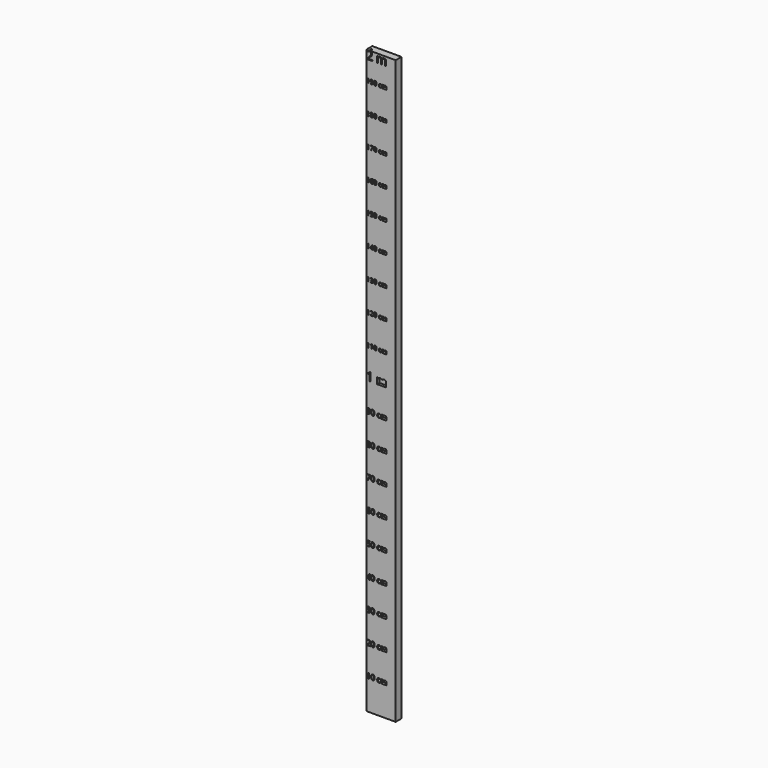
from build123d import *

# Parameters (mm, degrees)
F0_W         = 100
F0_H         = 2000
F1_DEPTH     = 25
F2_TEXT_SIZE = 40.1038403008
F3_DEPTH     = 10


# Not quite as in the source:
# - Text() gives the source's letters only with a copy of the font that has no kerning and outlines rounded to 1/6400 em; it was checked with that copy


with BuildPart() as f1:
    # F0 (on Front) → F1 (new body)
    with BuildSketch(Plane.XZ):
        with Locations((-11.6639206186, 561.5018179632)):
            Rectangle(F0_W, F0_H)
    extrude(amount=F1_DEPTH)

    # F2 (on face) → F3 (cut)
    with BuildSketch(Plane.XZ.offset(25)):
        with BuildLine():
            Line((-54.897684673, -325.7488393059), (-54.897684673, -338.4981820368))
            Line((-54.897684673, -338.4981820368), (-52.9163678972, -338.4981820368))
            Line((-52.9163678972, -338.4981820368), (-52.9163678972, -320.6075963681))
            Line((-52.9163678972, -320.6075963681), (-54.6275051126, -320.6075963681))
            Line((-54.6275051126, -320.6075963681), (-59.3615208871, -324.2687251928))
            Line((-59.3615208871, -324.2687251928), (-58.2847182916, -325.6626950983))
            add(Edge.make_bspline(
                [(-55.3734356379, -323.276108982), (-55.6925607707, -323.5560776569), (-58.2847182916, -325.6626950983)],
                knots=[0, 0, 0, 1, 1, 1], degree=2))
            add(Edge.make_bspline(
                [(-54.7997935279, -322.7377076843), (-55.054310505, -322.9961403072), (-55.3734356379, -323.276108982)],
                knots=[0, 0, 0, 1, 1, 1], degree=2))
            add(Edge.make_bspline(
                [(-54.897684673, -325.7488393059), (-54.897684673, -324.1551714646), (-54.7997935279, -322.7377076843)],
                knots=[0, 0, 0, 1, 1, 1], degree=2))
        make_face()
        with BuildLine():
            Line((-12.4129277227, -325.0870951654), (-12.4129277227, -338.4981820368))
            Line((-12.4129277227, -338.4981820368), (-10.3807075515, -338.4981820368))
            Line((-10.3807075515, -338.4981820368), (-10.3807075515, -331.4617665308))
            add(Edge.make_bspline(
                [(-9.4938137774, -327.7105778526), (-10.3807075515, -328.8539464268), (-10.3807075515, -331.4617665308)],
                knots=[0, 0, 0, 1, 1, 1], degree=2))
            add(Edge.make_bspline(
                [(-6.7000004978, -326.5672092785), (-8.6069200033, -326.5672092785), (-9.4938137774, -327.7105778526)],
                knots=[0, 0, 0, 1, 1, 1], degree=2))
            add(Edge.make_bspline(
                [(-4.5581422441, -327.367958845), (-5.2433802595, -326.5672092785), (-6.7000004978, -326.5672092785)],
                knots=[0, 0, 0, 1, 1, 1], degree=2))
            add(Edge.make_bspline(
                [(-3.8729042288, -329.7741231902), (-3.8729042288, -328.1687084115), (-4.5581422441, -327.367958845)],
                knots=[0, 0, 0, 1, 1, 1], degree=2))
            Line((-3.8729042288, -329.7741231902), (-3.8729042288, -338.4981820368))
            Line((-3.8729042288, -338.4981820368), (-1.8406840576, -338.4981820368))
            Line((-1.8406840576, -338.4981820368), (-1.8406840576, -331.0075516178))
            add(Edge.make_bspline(
                [(-0.9342120545, -327.6557588114), (-1.8406840576, -328.7443083443), (-1.8406840576, -331.0075516178)],
                knots=[0, 0, 0, 1, 1, 1], degree=2))
            add(Edge.make_bspline(
                [(1.8674325167, -326.5672092785), (-0.0277400514, -326.5672092785), (-0.9342120545, -327.6557588114)],
                knots=[0, 0, 0, 1, 1, 1], degree=2))
            add(Edge.make_bspline(
                [(3.9975438329, -327.367958845), (3.3123058176, -326.5672092785), (1.8674325167, -326.5672092785)],
                knots=[0, 0, 0, 1, 1, 1], degree=2))
            add(Edge.make_bspline(
                [(4.6827818483, -329.7741231902), (4.6827818483, -328.1687084115), (3.9975438329, -327.367958845)],
                knots=[0, 0, 0, 1, 1, 1], degree=2))
            Line((4.6827818483, -329.7741231902), (4.6827818483, -338.4981820368))
            Line((4.6827818483, -338.4981820368), (6.7110863736, -338.4981820368))
            Line((6.7110863736, -338.4981820368), (6.7110863736, -329.7506293154))
            add(Edge.make_bspline(
                [(5.5794647369, -326.0092297517), (6.7110863736, -327.1780500236), (6.7110863736, -329.7506293154)],
                knots=[0, 0, 0, 1, 1, 1], degree=2))
            add(Edge.make_bspline(
                [(2.1728528893, -324.8404094799), (4.4478431002, -324.8404094799), (5.5794647369, -326.0092297517)],
                knots=[0, 0, 0, 1, 1, 1], degree=2))
            add(Edge.make_bspline(
                [(-0.4212624545, -325.4532080479), (0.716232651, -324.8404094799), (2.1728528893, -324.8404094799)],
                knots=[0, 0, 0, 1, 1, 1], degree=2))
            add(Edge.make_bspline(
                [(-2.1578513676, -327.1193153366), (-1.5587575599, -326.0660066159), (-0.4212624545, -325.4532080479)],
                knots=[0, 0, 0, 1, 1, 1], degree=2))
            Line((-2.1578513676, -327.1193153366), (-2.2557425126, -327.1193153366))
            add(Edge.make_bspline(
                [(-6.3671706046, -324.8404094799), (-3.2229070257, -324.8404094799), (-2.2557425126, -327.1193153366)],
                knots=[0, 0, 0, 1, 1, 1], degree=2))
            add(Edge.make_bspline(
                [(-8.710684617, -325.3925155379), (-7.663249365, -324.8404094799), (-6.3671706046, -324.8404094799)],
                knots=[0, 0, 0, 1, 1, 1], degree=2))
            add(Edge.make_bspline(
                [(-10.3337198019, -326.9235330465), (-9.758119869, -325.944621596), (-8.710684617, -325.3925155379)],
                knots=[0, 0, 0, 1, 1, 1], degree=2))
            Line((-10.3337198019, -326.9235330465), (-10.4316109469, -326.9235330465))
            Line((-10.4316109469, -326.9235330465), (-10.7605251943, -325.0870951654))
            Line((-10.7605251943, -325.0870951654), (-12.4129277227, -325.0870951654))
        make_face()
        with BuildLine():
            add(Edge.make_bspline(
                [(-20.96335249, -338.4981820368), (-22.4891392415, -338.0797379108), (-23.494205342, -336.9515019451)],
                knots=[0.3708835197, 0.3708835197, 0.3708835197, 1, 1, 1], degree=2))
            Line((-20.96335249, -338.4981820368), (-16.8048665153, -338.4981820368))
            add(Edge.make_bspline(
                [(-15.5963477596, -338.0439671238), (-16.142629032, -338.3290526858), (-16.8048665153, -338.4981820368)],
                knots=[0, 0, 0, 0.406741787, 0.406741787, 0.406741787], degree=2))
            Line((-15.5963477596, -338.0439671238), (-15.5963477596, -336.2466857007))
            add(Edge.make_bspline(
                [(-19.0342847737, -336.9671645283), (-17.3583883705, -336.9671645283), (-15.5963477596, -336.2466857007)],
                knots=[0, 0, 0, 1, 1, 1], degree=2))
            add(Edge.make_bspline(
                [(-21.9886395312, -335.6456340701), (-20.9921076746, -336.9671645283), (-19.0342847737, -336.9671645283)],
                knots=[0, 0, 0, 1, 1, 1], degree=2))
            add(Edge.make_bspline(
                [(-22.9851713877, -331.853331111), (-22.9851713877, -334.324103612), (-21.9886395312, -335.6456340701)],
                knots=[0, 0, 0, 1, 1, 1], degree=2))
            add(Edge.make_bspline(
                [(-18.8972371706, -326.6416065487), (-22.9851713877, -326.6416065487), (-22.9851713877, -331.853331111)],
                knots=[0, 0, 0, 1, 1, 1], degree=2))
            add(Edge.make_bspline(
                [(-17.4915203277, -326.8178106098), (-18.2863964255, -326.6416065487), (-18.8972371706, -326.6416065487)],
                knots=[0, 0, 0, 1, 1, 1], degree=2))
            add(Edge.make_bspline(
                [(-16.023153152, -327.2641942312), (-16.6966442299, -326.9940146709), (-17.4915203277, -326.8178106098)],
                knots=[0, 0, 0, 1, 1, 1], degree=2))
            Line((-16.023153152, -327.2641942312), (-15.4005654695, -325.5413100784))
            add(Edge.make_bspline(
                [(-16.9159203948, -325.0498965303), (-15.9487558818, -325.2593835807), (-15.4005654695, -325.5413100784)],
                knots=[0, 0, 0, 1, 1, 1], degree=2))
            add(Edge.make_bspline(
                [(-18.850249421, -324.8404094799), (-17.8830849079, -324.8404094799), (-16.9159203948, -325.0498965303)],
                knots=[0, 0, 0, 1, 1, 1], degree=2))
            add(Edge.make_bspline(
                [(-23.4687536443, -326.676847361), (-21.8457184594, -324.8404094799), (-18.850249421, -324.8404094799)],
                knots=[0, 0, 0, 1, 1, 1], degree=2))
            add(Edge.make_bspline(
                [(-25.0917888291, -331.8768249858), (-25.0917888291, -328.513285242), (-23.4687536443, -326.676847361)],
                knots=[0, 0, 0, 1, 1, 1], degree=2))
            add(Edge.make_bspline(
                [(-23.494205342, -336.9515019451), (-25.0917888291, -335.1581361678), (-25.0917888291, -331.8768249858)],
                knots=[0, 0, 0, 1, 1, 1], degree=2))
        make_face()
        with BuildLine():
            Line((-16.8048665153, -338.4981820368), (-20.96335249, -338.4981820368))
            add(Edge.make_bspline(
                [(-18.9833813782, -338.7448677223), (-20.0638542598, -338.7448677223), (-20.96335249, -338.4981820368)],
                knots=[0, 0, 0, 0.3708835197, 0.3708835197, 0.3708835197], degree=2))
            add(Edge.make_bspline(
                [(-16.8048665153, -338.4981820368), (-17.770781104, -338.7448677223), (-18.9833813782, -338.7448677223)],
                knots=[0.406741787, 0.406741787, 0.406741787, 1, 1, 1], degree=2))
        make_face()
        with BuildLine():
            add(Edge.make_bspline(
                [(-41.9178023685, -338.4981820368), (-43.564820048, -337.9845313752), (-44.5819158079, -336.4013537099)],
                knots=[0.3244428423, 0.3244428423, 0.3244428423, 1, 1, 1], degree=2))
            Line((-41.9178023685, -338.4981820368), (-38.3802965964, -338.4981820368))
            add(Edge.make_bspline(
                [(-35.7168937125, -336.4561727511), (-36.6992428481, -337.9934768201), (-38.3802965964, -338.4981820368)],
                knots=[0, 0, 0, 0.6716946069, 0.6716946069, 0.6716946069], degree=2))
            add(Edge.make_bspline(
                [(-34.2544000055, -329.5274375047), (-34.2544000055, -334.1674777799), (-35.7168937125, -336.4561727511)],
                knots=[0, 0, 0, 1, 1, 1], degree=2))
            add(Edge.make_bspline(
                [(-35.765839285, -322.6887621118), (-34.2544000055, -325.0518543532), (-34.2544000055, -329.5274375047)],
                knots=[0, 0, 0, 1, 1, 1], degree=2))
            add(Edge.make_bspline(
                [(-40.1905190411, -320.3256698703), (-37.2772785646, -320.3256698703), (-35.765839285, -322.6887621118)],
                knots=[0, 0, 0, 1, 1, 1], degree=2))
            add(Edge.make_bspline(
                [(-44.6308613805, -322.5908709667), (-43.1742411422, -320.3256698703), (-40.1905190411, -320.3256698703)],
                knots=[0, 0, 0, 1, 1, 1], degree=2))
            add(Edge.make_bspline(
                [(-46.0874816188, -329.5274375047), (-46.0874816188, -324.8560720631), (-44.6308613805, -322.5908709667)],
                knots=[0, 0, 0, 1, 1, 1], degree=2))
            add(Edge.make_bspline(
                [(-44.5819158079, -336.4013537099), (-46.0874816188, -334.0578396975), (-46.0874816188, -329.5274375047)],
                knots=[0, 0, 0, 1, 1, 1], degree=2))
        make_face()
        with BuildLine():
            add(Edge.make_bspline(
                [(-44.0317675728, -329.5274375047), (-44.0317675728, -333.4313363692), (-43.1135486322, -335.212955209)],
                knots=[0, 0, 0, 1, 1, 1], degree=2))
            add(Edge.make_bspline(
                [(-43.1135486322, -323.8556245607), (-44.0317675728, -325.6235386403), (-44.0317675728, -329.5274375047)],
                knots=[0, 0, 0, 1, 1, 1], degree=2))
            add(Edge.make_bspline(
                [(-40.1905190411, -322.0877104812), (-42.1953296917, -322.0877104812), (-43.1135486322, -323.8556245607)],
                knots=[0, 0, 0, 1, 1, 1], degree=2))
            add(Edge.make_bspline(
                [(-37.247911221, -323.8810762584), (-38.15829887, -322.0877104812), (-40.1905190411, -322.0877104812)],
                knots=[0, 0, 0, 1, 1, 1], degree=2))
            add(Edge.make_bspline(
                [(-36.3375235721, -329.5274375047), (-36.3375235721, -325.6744420357), (-37.247911221, -323.8810762584)],
                knots=[0, 0, 0, 1, 1, 1], degree=2))
            add(Edge.make_bspline(
                [(-37.247911221, -335.1894613342), (-36.3375235721, -333.3843486196), (-36.3375235721, -329.5274375047)],
                knots=[0, 0, 0, 1, 1, 1], degree=2))
            add(Edge.make_bspline(
                [(-40.1905190411, -336.9945740489), (-38.15829887, -336.9945740489), (-37.247911221, -335.1894613342)],
                knots=[0, 0, 0, 1, 1, 1], degree=2))
            add(Edge.make_bspline(
                [(-43.1135486322, -335.212955209), (-42.1953296917, -336.9945740489), (-40.1905190411, -336.9945740489)],
                knots=[0, 0, 0, 1, 1, 1], degree=2))
        make_face(mode=Mode.SUBTRACT)
        with BuildLine():
            Line((-38.3802965964, -338.4981820368), (-41.9178023685, -338.4981820368))
            add(Edge.make_bspline(
                [(-40.1905190411, -338.7448677223), (-41.1268062388, -338.7448677223), (-41.9178023685, -338.4981820368)],
                knots=[0, 0, 0, 0.3244428423, 0.3244428423, 0.3244428423], degree=2))
            add(Edge.make_bspline(
                [(-38.3802965964, -338.4981820368), (-39.2019482904, -338.7448677223), (-40.1905190411, -338.7448677223)],
                knots=[0.6716946069, 0.6716946069, 0.6716946069, 1, 1, 1], degree=2))
        make_face()
        with BuildLine():
            Line((-10.3807075515, -331.4617665308), (-10.3807075515, -338.4981820368))
            Line((-10.3807075515, -338.4981820368), (-3.8729042288, -338.4981820368))
            Line((-3.8729042288, -338.4981820368), (-3.8729042288, -329.7741231902))
            add(Edge.make_bspline(
                [(-3.8729042288, -329.7741231902), (-3.8729042288, -328.1687084115), (-4.5581422441, -327.367958845)],
                knots=[0, 0, 0, 1, 1, 1], degree=2))
            add(Edge.make_bspline(
                [(-4.5581422441, -327.367958845), (-5.2433802595, -326.5672092785), (-6.7000004978, -326.5672092785)],
                knots=[0, 0, 0, 1, 1, 1], degree=2))
            add(Edge.make_bspline(
                [(-6.7000004978, -326.5672092785), (-8.6069200033, -326.5672092785), (-9.4938137774, -327.7105778526)],
                knots=[0, 0, 0, 1, 1, 1], degree=2))
            add(Edge.make_bspline(
                [(-9.4938137774, -327.7105778526), (-10.3807075515, -328.8539464268), (-10.3807075515, -331.4617665308)],
                knots=[0, 0, 0, 1, 1, 1], degree=2))
        make_face()
        with BuildLine():
            Line((-1.8406840576, -331.0075516178), (-1.8406840576, -338.4981820368))
            Line((-1.8406840576, -338.4981820368), (4.6827818483, -338.4981820368))
            Line((4.6827818483, -338.4981820368), (4.6827818483, -329.7741231902))
            add(Edge.make_bspline(
                [(4.6827818483, -329.7741231902), (4.6827818483, -328.1687084115), (3.9975438329, -327.367958845)],
                knots=[0, 0, 0, 1, 1, 1], degree=2))
            add(Edge.make_bspline(
                [(3.9975438329, -327.367958845), (3.3123058176, -326.5672092785), (1.8674325167, -326.5672092785)],
                knots=[0, 0, 0, 1, 1, 1], degree=2))
            add(Edge.make_bspline(
                [(1.8674325167, -326.5672092785), (-0.0277400514, -326.5672092785), (-0.9342120545, -327.6557588114)],
                knots=[0, 0, 0, 1, 1, 1], degree=2))
            add(Edge.make_bspline(
                [(-0.9342120545, -327.6557588114), (-1.8406840576, -328.7443083443), (-1.8406840576, -331.0075516178)],
                knots=[0, 0, 0, 1, 1, 1], degree=2))
        make_face()
        with BuildLine():
            Line((-60.4383234826, -236.7478883634), (-60.4383234826, -238.4981820368))
            Line((-60.4383234826, -238.4981820368), (-48.6796391396, -238.4981820368))
            Line((-48.6796391396, -238.4981820368), (-48.6796391396, -236.6147564061))
            Line((-48.6796391396, -236.6147564061), (-57.881406774, -236.6147564061))
            Line((-57.881406774, -236.6147564061), (-57.881406774, -236.516865261))
            Line((-57.881406774, -236.516865261), (-53.9657609721, -232.6873636668))
            add(Edge.make_bspline(
                [(-50.3946920008, -228.4780444298), (-51.3501095765, -230.1421938956), (-53.9657609721, -232.6873636668)],
                knots=[0, 0, 0, 1, 1, 1], degree=2))
            add(Edge.make_bspline(
                [(-49.4392744252, -225.1105890402), (-49.4392744252, -226.813894964), (-50.3946920008, -228.4780444298)],
                knots=[0, 0, 0, 1, 1, 1], degree=2))
            add(Edge.make_bspline(
                [(-50.8704429657, -221.6432846827), (-49.4392744252, -222.9334899744), (-49.4392744252, -225.1105890402)],
                knots=[0, 0, 0, 1, 1, 1], degree=2))
            add(Edge.make_bspline(
                [(-54.8232874027, -220.3530793909), (-52.3016115063, -220.3530793909), (-50.8704429657, -221.6432846827)],
                knots=[0, 0, 0, 1, 1, 1], degree=2))
            add(Edge.make_bspline(
                [(-60.2073003803, -222.4087934369), (-57.7365278793, -220.3530793909), (-54.8232874027, -220.3530793909)],
                knots=[0, 0, 0, 1, 1, 1], degree=2))
            Line((-60.2073003803, -222.4087934369), (-59.1304977848, -223.791016405))
            add(Edge.make_bspline(
                [(-56.9103266151, -222.4557811865), (-57.9088162946, -222.8238518919), (-59.1304977848, -223.791016405)],
                knots=[0, 0, 0, 1, 1, 1], degree=2))
            add(Edge.make_bspline(
                [(-54.7997935279, -222.0877104812), (-55.9118369356, -222.0877104812), (-56.9103266151, -222.4557811865)],
                knots=[0, 0, 0, 1, 1, 1], degree=2))
            add(Edge.make_bspline(
                [(-52.387755714, -222.9256586828), (-53.257029082, -222.0877104812), (-54.7997935279, -222.0877104812)],
                knots=[0, 0, 0, 1, 1, 1], degree=2))
            add(Edge.make_bspline(
                [(-51.518482346, -225.1967332478), (-51.518482346, -223.7636068844), (-52.387755714, -222.9256586828)],
                knots=[0, 0, 0, 1, 1, 1], degree=2))
            add(Edge.make_bspline(
                [(-51.8611013536, -227.091905816), (-51.518482346, -226.2108855105), (-51.518482346, -225.1967332478)],
                knots=[0, 0, 0, 1, 1, 1], degree=2))
            add(Edge.make_bspline(
                [(-52.8889583766, -228.9028919993), (-52.2037203613, -227.9729261214), (-51.8611013536, -227.091905816)],
                knots=[0, 0, 0, 1, 1, 1], degree=2))
            add(Edge.make_bspline(
                [(-55.727801583, -232.0138725889), (-53.5741963919, -229.8328578773), (-52.8889583766, -228.9028919993)],
                knots=[0, 0, 0, 1, 1, 1], degree=2))
            Line((-55.727801583, -232.0138725889), (-60.4383234826, -236.7478883634))
        make_face()
        with BuildLine():
            Line((-12.4129277227, -225.0870951654), (-12.4129277227, -238.4981820368))
            Line((-12.4129277227, -238.4981820368), (-10.3807075515, -238.4981820368))
            Line((-10.3807075515, -238.4981820368), (-10.3807075515, -231.4617665308))
            add(Edge.make_bspline(
                [(-9.4938137774, -227.7105778526), (-10.3807075515, -228.8539464268), (-10.3807075515, -231.4617665308)],
                knots=[0, 0, 0, 1, 1, 1], degree=2))
            add(Edge.make_bspline(
                [(-6.7000004978, -226.5672092785), (-8.6069200033, -226.5672092785), (-9.4938137774, -227.7105778526)],
                knots=[0, 0, 0, 1, 1, 1], degree=2))
            add(Edge.make_bspline(
                [(-4.5581422441, -227.367958845), (-5.2433802595, -226.5672092785), (-6.7000004978, -226.5672092785)],
                knots=[0, 0, 0, 1, 1, 1], degree=2))
            add(Edge.make_bspline(
                [(-3.8729042288, -229.7741231902), (-3.8729042288, -228.1687084115), (-4.5581422441, -227.367958845)],
                knots=[0, 0, 0, 1, 1, 1], degree=2))
            Line((-3.8729042288, -229.7741231902), (-3.8729042288, -238.4981820368))
            Line((-3.8729042288, -238.4981820368), (-1.8406840576, -238.4981820368))
            Line((-1.8406840576, -238.4981820368), (-1.8406840576, -231.0075516178))
            add(Edge.make_bspline(
                [(-0.9342120545, -227.6557588114), (-1.8406840576, -228.7443083443), (-1.8406840576, -231.0075516178)],
                knots=[0, 0, 0, 1, 1, 1], degree=2))
            add(Edge.make_bspline(
                [(1.8674325167, -226.5672092785), (-0.0277400514, -226.5672092785), (-0.9342120545, -227.6557588114)],
                knots=[0, 0, 0, 1, 1, 1], degree=2))
            add(Edge.make_bspline(
                [(3.9975438329, -227.367958845), (3.3123058176, -226.5672092785), (1.8674325167, -226.5672092785)],
                knots=[0, 0, 0, 1, 1, 1], degree=2))
            add(Edge.make_bspline(
                [(4.6827818483, -229.7741231902), (4.6827818483, -228.1687084115), (3.9975438329, -227.367958845)],
                knots=[0, 0, 0, 1, 1, 1], degree=2))
            Line((4.6827818483, -229.7741231902), (4.6827818483, -238.4981820368))
            Line((4.6827818483, -238.4981820368), (6.7110863736, -238.4981820368))
            Line((6.7110863736, -238.4981820368), (6.7110863736, -229.7506293154))
            add(Edge.make_bspline(
                [(5.5794647369, -226.0092297517), (6.7110863736, -227.1780500236), (6.7110863736, -229.7506293154)],
                knots=[0, 0, 0, 1, 1, 1], degree=2))
            add(Edge.make_bspline(
                [(2.1728528893, -224.8404094799), (4.4478431002, -224.8404094799), (5.5794647369, -226.0092297517)],
                knots=[0, 0, 0, 1, 1, 1], degree=2))
            add(Edge.make_bspline(
                [(-0.4212624545, -225.4532080479), (0.716232651, -224.8404094799), (2.1728528893, -224.8404094799)],
                knots=[0, 0, 0, 1, 1, 1], degree=2))
            add(Edge.make_bspline(
                [(-2.1578513676, -227.1193153366), (-1.5587575599, -226.0660066159), (-0.4212624545, -225.4532080479)],
                knots=[0, 0, 0, 1, 1, 1], degree=2))
            Line((-2.1578513676, -227.1193153366), (-2.2557425126, -227.1193153366))
            add(Edge.make_bspline(
                [(-6.3671706046, -224.8404094799), (-3.2229070257, -224.8404094799), (-2.2557425126, -227.1193153366)],
                knots=[0, 0, 0, 1, 1, 1], degree=2))
            add(Edge.make_bspline(
                [(-8.710684617, -225.3925155379), (-7.663249365, -224.8404094799), (-6.3671706046, -224.8404094799)],
                knots=[0, 0, 0, 1, 1, 1], degree=2))
            add(Edge.make_bspline(
                [(-10.3337198019, -226.9235330465), (-9.758119869, -225.944621596), (-8.710684617, -225.3925155379)],
                knots=[0, 0, 0, 1, 1, 1], degree=2))
            Line((-10.3337198019, -226.9235330465), (-10.4316109469, -226.9235330465))
            Line((-10.4316109469, -226.9235330465), (-10.7605251943, -225.0870951654))
            Line((-10.7605251943, -225.0870951654), (-12.4129277227, -225.0870951654))
        make_face()
        with BuildLine():
            add(Edge.make_bspline(
                [(-20.96335249, -238.4981820368), (-22.4891392415, -238.0797379108), (-23.494205342, -236.9515019451)],
                knots=[0.3708835197, 0.3708835197, 0.3708835197, 1, 1, 1], degree=2))
            Line((-20.96335249, -238.4981820368), (-16.8048665153, -238.4981820368))
            add(Edge.make_bspline(
                [(-15.5963477596, -238.0439671238), (-16.142629032, -238.3290526858), (-16.8048665153, -238.4981820368)],
                knots=[0, 0, 0, 0.406741787, 0.406741787, 0.406741787], degree=2))
            Line((-15.5963477596, -238.0439671238), (-15.5963477596, -236.2466857007))
            add(Edge.make_bspline(
                [(-19.0342847737, -236.9671645283), (-17.3583883705, -236.9671645283), (-15.5963477596, -236.2466857007)],
                knots=[0, 0, 0, 1, 1, 1], degree=2))
            add(Edge.make_bspline(
                [(-21.9886395312, -235.6456340701), (-20.9921076746, -236.9671645283), (-19.0342847737, -236.9671645283)],
                knots=[0, 0, 0, 1, 1, 1], degree=2))
            add(Edge.make_bspline(
                [(-22.9851713877, -231.853331111), (-22.9851713877, -234.324103612), (-21.9886395312, -235.6456340701)],
                knots=[0, 0, 0, 1, 1, 1], degree=2))
            add(Edge.make_bspline(
                [(-18.8972371706, -226.6416065487), (-22.9851713877, -226.6416065487), (-22.9851713877, -231.853331111)],
                knots=[0, 0, 0, 1, 1, 1], degree=2))
            add(Edge.make_bspline(
                [(-17.4915203277, -226.8178106098), (-18.2863964255, -226.6416065487), (-18.8972371706, -226.6416065487)],
                knots=[0, 0, 0, 1, 1, 1], degree=2))
            add(Edge.make_bspline(
                [(-16.023153152, -227.2641942312), (-16.6966442299, -226.9940146709), (-17.4915203277, -226.8178106098)],
                knots=[0, 0, 0, 1, 1, 1], degree=2))
            Line((-16.023153152, -227.2641942312), (-15.4005654695, -225.5413100784))
            add(Edge.make_bspline(
                [(-16.9159203948, -225.0498965303), (-15.9487558818, -225.2593835807), (-15.4005654695, -225.5413100784)],
                knots=[0, 0, 0, 1, 1, 1], degree=2))
            add(Edge.make_bspline(
                [(-18.850249421, -224.8404094799), (-17.8830849079, -224.8404094799), (-16.9159203948, -225.0498965303)],
                knots=[0, 0, 0, 1, 1, 1], degree=2))
            add(Edge.make_bspline(
                [(-23.4687536443, -226.676847361), (-21.8457184594, -224.8404094799), (-18.850249421, -224.8404094799)],
                knots=[0, 0, 0, 1, 1, 1], degree=2))
            add(Edge.make_bspline(
                [(-25.0917888291, -231.8768249858), (-25.0917888291, -228.513285242), (-23.4687536443, -226.676847361)],
                knots=[0, 0, 0, 1, 1, 1], degree=2))
            add(Edge.make_bspline(
                [(-23.494205342, -236.9515019451), (-25.0917888291, -235.1581361678), (-25.0917888291, -231.8768249858)],
                knots=[0, 0, 0, 1, 1, 1], degree=2))
        make_face()
        with BuildLine():
            Line((-16.8048665153, -238.4981820368), (-20.96335249, -238.4981820368))
            add(Edge.make_bspline(
                [(-18.9833813782, -238.7448677223), (-20.0638542598, -238.7448677223), (-20.96335249, -238.4981820368)],
                knots=[0, 0, 0, 0.3708835197, 0.3708835197, 0.3708835197], degree=2))
            add(Edge.make_bspline(
                [(-16.8048665153, -238.4981820368), (-17.770781104, -238.7448677223), (-18.9833813782, -238.7448677223)],
                knots=[0.406741787, 0.406741787, 0.406741787, 1, 1, 1], degree=2))
        make_face()
        with BuildLine():
            add(Edge.make_bspline(
                [(-41.9178023685, -238.4981820368), (-43.564820048, -237.9845313752), (-44.5819158079, -236.4013537099)],
                knots=[0.3244428423, 0.3244428423, 0.3244428423, 1, 1, 1], degree=2))
            Line((-41.9178023685, -238.4981820368), (-38.3802965964, -238.4981820368))
            add(Edge.make_bspline(
                [(-35.7168937125, -236.4561727511), (-36.6992428481, -237.9934768201), (-38.3802965964, -238.4981820368)],
                knots=[0, 0, 0, 0.6716946069, 0.6716946069, 0.6716946069], degree=2))
            add(Edge.make_bspline(
                [(-34.2544000055, -229.5274375047), (-34.2544000055, -234.1674777799), (-35.7168937125, -236.4561727511)],
                knots=[0, 0, 0, 1, 1, 1], degree=2))
            add(Edge.make_bspline(
                [(-35.765839285, -222.6887621118), (-34.2544000055, -225.0518543532), (-34.2544000055, -229.5274375047)],
                knots=[0, 0, 0, 1, 1, 1], degree=2))
            add(Edge.make_bspline(
                [(-40.1905190411, -220.3256698703), (-37.2772785646, -220.3256698703), (-35.765839285, -222.6887621118)],
                knots=[0, 0, 0, 1, 1, 1], degree=2))
            add(Edge.make_bspline(
                [(-44.6308613805, -222.5908709667), (-43.1742411422, -220.3256698703), (-40.1905190411, -220.3256698703)],
                knots=[0, 0, 0, 1, 1, 1], degree=2))
            add(Edge.make_bspline(
                [(-46.0874816188, -229.5274375047), (-46.0874816188, -224.8560720631), (-44.6308613805, -222.5908709667)],
                knots=[0, 0, 0, 1, 1, 1], degree=2))
            add(Edge.make_bspline(
                [(-44.5819158079, -236.4013537099), (-46.0874816188, -234.0578396975), (-46.0874816188, -229.5274375047)],
                knots=[0, 0, 0, 1, 1, 1], degree=2))
        make_face()
        with BuildLine():
            add(Edge.make_bspline(
                [(-44.0317675728, -229.5274375047), (-44.0317675728, -233.4313363692), (-43.1135486322, -235.212955209)],
                knots=[0, 0, 0, 1, 1, 1], degree=2))
            add(Edge.make_bspline(
                [(-43.1135486322, -223.8556245607), (-44.0317675728, -225.6235386403), (-44.0317675728, -229.5274375047)],
                knots=[0, 0, 0, 1, 1, 1], degree=2))
            add(Edge.make_bspline(
                [(-40.1905190411, -222.0877104812), (-42.1953296917, -222.0877104812), (-43.1135486322, -223.8556245607)],
                knots=[0, 0, 0, 1, 1, 1], degree=2))
            add(Edge.make_bspline(
                [(-37.247911221, -223.8810762584), (-38.15829887, -222.0877104812), (-40.1905190411, -222.0877104812)],
                knots=[0, 0, 0, 1, 1, 1], degree=2))
            add(Edge.make_bspline(
                [(-36.3375235721, -229.5274375047), (-36.3375235721, -225.6744420357), (-37.247911221, -223.8810762584)],
                knots=[0, 0, 0, 1, 1, 1], degree=2))
            add(Edge.make_bspline(
                [(-37.247911221, -235.1894613342), (-36.3375235721, -233.3843486196), (-36.3375235721, -229.5274375047)],
                knots=[0, 0, 0, 1, 1, 1], degree=2))
            add(Edge.make_bspline(
                [(-40.1905190411, -236.9945740489), (-38.15829887, -236.9945740489), (-37.247911221, -235.1894613342)],
                knots=[0, 0, 0, 1, 1, 1], degree=2))
            add(Edge.make_bspline(
                [(-43.1135486322, -235.212955209), (-42.1953296917, -236.9945740489), (-40.1905190411, -236.9945740489)],
                knots=[0, 0, 0, 1, 1, 1], degree=2))
        make_face(mode=Mode.SUBTRACT)
        with BuildLine():
            Line((-38.3802965964, -238.4981820368), (-41.9178023685, -238.4981820368))
            add(Edge.make_bspline(
                [(-40.1905190411, -238.7448677223), (-41.1268062388, -238.7448677223), (-41.9178023685, -238.4981820368)],
                knots=[0, 0, 0, 0.3244428423, 0.3244428423, 0.3244428423], degree=2))
            add(Edge.make_bspline(
                [(-38.3802965964, -238.4981820368), (-39.2019482904, -238.7448677223), (-40.1905190411, -238.7448677223)],
                knots=[0.6716946069, 0.6716946069, 0.6716946069, 1, 1, 1], degree=2))
        make_face()
        with BuildLine():
            Line((-10.3807075515, -231.4617665308), (-10.3807075515, -238.4981820368))
            Line((-10.3807075515, -238.4981820368), (-3.8729042288, -238.4981820368))
            Line((-3.8729042288, -238.4981820368), (-3.8729042288, -229.7741231902))
            add(Edge.make_bspline(
                [(-3.8729042288, -229.7741231902), (-3.8729042288, -228.1687084115), (-4.5581422441, -227.367958845)],
                knots=[0, 0, 0, 1, 1, 1], degree=2))
            add(Edge.make_bspline(
                [(-4.5581422441, -227.367958845), (-5.2433802595, -226.5672092785), (-6.7000004978, -226.5672092785)],
                knots=[0, 0, 0, 1, 1, 1], degree=2))
            add(Edge.make_bspline(
                [(-6.7000004978, -226.5672092785), (-8.6069200033, -226.5672092785), (-9.4938137774, -227.7105778526)],
                knots=[0, 0, 0, 1, 1, 1], degree=2))
            add(Edge.make_bspline(
                [(-9.4938137774, -227.7105778526), (-10.3807075515, -228.8539464268), (-10.3807075515, -231.4617665308)],
                knots=[0, 0, 0, 1, 1, 1], degree=2))
        make_face()
        with BuildLine():
            Line((-1.8406840576, -231.0075516178), (-1.8406840576, -238.4981820368))
            Line((-1.8406840576, -238.4981820368), (4.6827818483, -238.4981820368))
            Line((4.6827818483, -238.4981820368), (4.6827818483, -229.7741231902))
            add(Edge.make_bspline(
                [(4.6827818483, -229.7741231902), (4.6827818483, -228.1687084115), (3.9975438329, -227.367958845)],
                knots=[0, 0, 0, 1, 1, 1], degree=2))
            add(Edge.make_bspline(
                [(3.9975438329, -227.367958845), (3.3123058176, -226.5672092785), (1.8674325167, -226.5672092785)],
                knots=[0, 0, 0, 1, 1, 1], degree=2))
            add(Edge.make_bspline(
                [(1.8674325167, -226.5672092785), (-0.0277400514, -226.5672092785), (-0.9342120545, -227.6557588114)],
                knots=[0, 0, 0, 1, 1, 1], degree=2))
            add(Edge.make_bspline(
                [(-0.9342120545, -227.6557588114), (-1.8406840576, -228.7443083443), (-1.8406840576, -231.0075516178)],
                knots=[0, 0, 0, 1, 1, 1], degree=2))
        make_face()
        with BuildLine():
            Line((-12.4129277227, -125.0870951654), (-12.4129277227, -138.4981820368))
            Line((-12.4129277227, -138.4981820368), (-10.3807075515, -138.4981820368))
            Line((-10.3807075515, -138.4981820368), (-10.3807075515, -131.4617665308))
            add(Edge.make_bspline(
                [(-9.4938137774, -127.7105778526), (-10.3807075515, -128.8539464268), (-10.3807075515, -131.4617665308)],
                knots=[0, 0, 0, 1, 1, 1], degree=2))
            add(Edge.make_bspline(
                [(-6.7000004978, -126.5672092785), (-8.6069200033, -126.5672092785), (-9.4938137774, -127.7105778526)],
                knots=[0, 0, 0, 1, 1, 1], degree=2))
            add(Edge.make_bspline(
                [(-4.5581422441, -127.367958845), (-5.2433802595, -126.5672092785), (-6.7000004978, -126.5672092785)],
                knots=[0, 0, 0, 1, 1, 1], degree=2))
            add(Edge.make_bspline(
                [(-3.8729042288, -129.7741231902), (-3.8729042288, -128.1687084115), (-4.5581422441, -127.367958845)],
                knots=[0, 0, 0, 1, 1, 1], degree=2))
            Line((-3.8729042288, -129.7741231902), (-3.8729042288, -138.4981820368))
            Line((-3.8729042288, -138.4981820368), (-1.8406840576, -138.4981820368))
            Line((-1.8406840576, -138.4981820368), (-1.8406840576, -131.0075516178))
            add(Edge.make_bspline(
                [(-0.9342120545, -127.6557588114), (-1.8406840576, -128.7443083443), (-1.8406840576, -131.0075516178)],
                knots=[0, 0, 0, 1, 1, 1], degree=2))
            add(Edge.make_bspline(
                [(1.8674325167, -126.5672092785), (-0.0277400514, -126.5672092785), (-0.9342120545, -127.6557588114)],
                knots=[0, 0, 0, 1, 1, 1], degree=2))
            add(Edge.make_bspline(
                [(3.9975438329, -127.367958845), (3.3123058176, -126.5672092785), (1.8674325167, -126.5672092785)],
                knots=[0, 0, 0, 1, 1, 1], degree=2))
            add(Edge.make_bspline(
                [(4.6827818483, -129.7741231902), (4.6827818483, -128.1687084115), (3.9975438329, -127.367958845)],
                knots=[0, 0, 0, 1, 1, 1], degree=2))
            Line((4.6827818483, -129.7741231902), (4.6827818483, -138.4981820368))
            Line((4.6827818483, -138.4981820368), (6.7110863736, -138.4981820368))
            Line((6.7110863736, -138.4981820368), (6.7110863736, -129.7506293154))
            add(Edge.make_bspline(
                [(5.5794647369, -126.0092297517), (6.7110863736, -127.1780500236), (6.7110863736, -129.7506293154)],
                knots=[0, 0, 0, 1, 1, 1], degree=2))
            add(Edge.make_bspline(
                [(2.1728528893, -124.8404094799), (4.4478431002, -124.8404094799), (5.5794647369, -126.0092297517)],
                knots=[0, 0, 0, 1, 1, 1], degree=2))
            add(Edge.make_bspline(
                [(-0.4212624545, -125.4532080479), (0.716232651, -124.8404094799), (2.1728528893, -124.8404094799)],
                knots=[0, 0, 0, 1, 1, 1], degree=2))
            add(Edge.make_bspline(
                [(-2.1578513676, -127.1193153366), (-1.5587575599, -126.0660066159), (-0.4212624545, -125.4532080479)],
                knots=[0, 0, 0, 1, 1, 1], degree=2))
            Line((-2.1578513676, -127.1193153366), (-2.2557425126, -127.1193153366))
            add(Edge.make_bspline(
                [(-6.3671706046, -124.8404094799), (-3.2229070257, -124.8404094799), (-2.2557425126, -127.1193153366)],
                knots=[0, 0, 0, 1, 1, 1], degree=2))
            add(Edge.make_bspline(
                [(-8.710684617, -125.3925155379), (-7.663249365, -124.8404094799), (-6.3671706046, -124.8404094799)],
                knots=[0, 0, 0, 1, 1, 1], degree=2))
            add(Edge.make_bspline(
                [(-10.3337198019, -126.9235330465), (-9.758119869, -125.944621596), (-8.710684617, -125.3925155379)],
                knots=[0, 0, 0, 1, 1, 1], degree=2))
            Line((-10.3337198019, -126.9235330465), (-10.4316109469, -126.9235330465))
            Line((-10.4316109469, -126.9235330465), (-10.7605251943, -125.0870951654))
            Line((-10.7605251943, -125.0870951654), (-12.4129277227, -125.0870951654))
        make_face()
        with BuildLine():
            add(Edge.make_bspline(
                [(-53.1220613576, -138.4981820368), (-54.236607818, -138.7448677223), (-55.6181635005, -138.7448677223)],
                knots=[0.5769429439, 0.5769429439, 0.5769429439, 1, 1, 1], degree=2))
            Line((-53.1220613576, -138.4981820368), (-58.3830820276, -138.4981820368))
            add(Edge.make_bspline(
                [(-58.2201101359, -138.5295072032), (-58.3017599673, -138.5146125408), (-58.3830820276, -138.4981820368)],
                knots=[0, 0, 0, 0.0691615274, 0.0691615274, 0.0691615274], degree=2))
            add(Edge.make_bspline(
                [(-55.6181635005, -138.7448677223), (-57.0395429266, -138.7448677223), (-58.2201101359, -138.5295072032)],
                knots=[0, 0, 0, 1, 1, 1], degree=2))
        make_face()
        with BuildLine():
            Line((-58.3830820276, -138.4981820368), (-53.1220613576, -138.4981820368))
            add(Edge.make_bspline(
                [(-50.5787273535, -137.3665604001), (-51.6021015634, -138.1617650841), (-53.1220613576, -138.4981820368)],
                knots=[0, 0, 0, 0.5769429439, 0.5769429439, 0.5769429439], degree=2))
            add(Edge.make_bspline(
                [(-48.8049398053, -133.4313363692), (-48.8049398053, -135.9882530778), (-50.5787273535, -137.3665604001)],
                knots=[0, 0, 0, 1, 1, 1], degree=2))
            add(Edge.make_bspline(
                [(-49.8445437657, -130.5435475903), (-48.8049398053, -131.6458018835), (-48.8049398053, -133.4313363692)],
                knots=[0, 0, 0, 1, 1, 1], degree=2))
            add(Edge.make_bspline(
                [(-53.0377529171, -129.1750293825), (-50.8841477261, -129.4412932971), (-49.8445437657, -130.5435475903)],
                knots=[0, 0, 0, 1, 1, 1], degree=2))
            Line((-53.0377529171, -129.1750293825), (-53.0377529171, -129.0771382375))
            add(Edge.make_bspline(
                [(-50.3144212619, -127.6205179992), (-51.2757123062, -128.7090675321), (-53.0377529171, -129.0771382375)],
                knots=[0, 0, 0, 1, 1, 1], degree=2))
            add(Edge.make_bspline(
                [(-49.3531302175, -124.8169156051), (-49.3531302175, -126.5319684663), (-50.3144212619, -127.6205179992)],
                knots=[0, 0, 0, 1, 1, 1], degree=2))
            add(Edge.make_bspline(
                [(-50.7980035184, -121.5453935376), (-49.3531302175, -122.7377076843), (-49.3531302175, -124.8169156051)],
                knots=[0, 0, 0, 1, 1, 1], degree=2))
            add(Edge.make_bspline(
                [(-54.8467812775, -120.3530793909), (-52.2428768193, -120.3530793909), (-50.7980035184, -121.5453935376)],
                knots=[0, 0, 0, 1, 1, 1], degree=2))
            add(Edge.make_bspline(
                [(-57.8774911282, -120.8484085849), (-56.4404491189, -120.3530793909), (-54.8467812775, -120.3530793909)],
                knots=[0, 0, 0, 1, 1, 1], degree=2))
            add(Edge.make_bspline(
                [(-60.4148296078, -122.2130111468), (-59.3145331375, -121.3437377788), (-57.8774911282, -120.8484085849)],
                knots=[0, 0, 0, 1, 1, 1], degree=2))
            Line((-60.4148296078, -122.2130111468), (-59.3889304077, -123.5834871775))
            add(Edge.make_bspline(
                [(-57.0140912289, -122.406835614), (-58.0536951893, -122.7259607469), (-59.3889304077, -123.5834871775)],
                knots=[0, 0, 0, 1, 1, 1], degree=2))
            add(Edge.make_bspline(
                [(-54.7997935279, -122.0877104812), (-55.9744872685, -122.0877104812), (-57.0140912289, -122.406835614)],
                knots=[0, 0, 0, 1, 1, 1], degree=2))
            add(Edge.make_bspline(
                [(-52.3583883705, -122.8355988293), (-53.257029082, -122.0877104812), (-54.7997935279, -122.0877104812)],
                knots=[0, 0, 0, 1, 1, 1], degree=2))
            add(Edge.make_bspline(
                [(-51.4597476589, -124.8913128753), (-51.4597476589, -123.5834871775), (-52.3583883705, -122.8355988293)],
                knots=[0, 0, 0, 1, 1, 1], degree=2))
            add(Edge.make_bspline(
                [(-52.683386972, -127.4560608755), (-51.4597476589, -126.5319684663), (-51.4597476589, -124.8913128753)],
                knots=[0, 0, 0, 1, 1, 1], degree=2))
            add(Edge.make_bspline(
                [(-55.9979811433, -128.3801532848), (-53.9070262851, -128.3801532848), (-52.683386972, -127.4560608755)],
                knots=[0, 0, 0, 1, 1, 1], degree=2))
            Line((-55.9979811433, -128.3801532848), (-57.7835156289, -128.3801532848))
            Line((-57.7835156289, -128.3801532848), (-57.7835156289, -130.1265313124))
            Line((-57.7835156289, -130.1265313124), (-56.0214750181, -130.1265313124))
            add(Edge.make_bspline(
                [(-50.9076416009, -133.3843486196), (-50.9076416009, -130.1265313124), (-56.0214750181, -130.1265313124)],
                knots=[0, 0, 0, 1, 1, 1], degree=2))
            add(Edge.make_bspline(
                [(-55.5437662303, -137.0180679237), (-50.9076416009, -137.0180679237), (-50.9076416009, -133.3843486196)],
                knots=[0, 0, 0, 1, 1, 1], degree=2))
            add(Edge.make_bspline(
                [(-58.0341169603, -136.7185210198), (-56.7184599708, -137.0180679237), (-55.5437662303, -137.0180679237)],
                knots=[0, 0, 0, 1, 1, 1], degree=2))
            add(Edge.make_bspline(
                [(-60.5127207528, -135.8433741831), (-59.3497739497, -136.418974116), (-58.0341169603, -136.7185210198)],
                knots=[0, 0, 0, 1, 1, 1], degree=2))
            Line((-60.5127207528, -135.8433741831), (-60.5127207528, -137.7777032093))
            add(Edge.make_bspline(
                [(-58.3830820276, -138.4981820368), (-59.4775879658, -138.277045434), (-60.5127207528, -137.7777032093)],
                knots=[0.0691615274, 0.0691615274, 0.0691615274, 1, 1, 1], degree=2))
        make_face()
        with BuildLine():
            add(Edge.make_bspline(
                [(-38.3802965964, -138.4981820368), (-39.2019482904, -138.7448677223), (-40.1905190411, -138.7448677223)],
                knots=[0.6716946069, 0.6716946069, 0.6716946069, 1, 1, 1], degree=2))
            Line((-38.3802965964, -138.4981820368), (-41.9178023685, -138.4981820368))
            add(Edge.make_bspline(
                [(-40.1905190411, -138.7448677223), (-41.1268062388, -138.7448677223), (-41.9178023685, -138.4981820368)],
                knots=[0, 0, 0, 0.3244428423, 0.3244428423, 0.3244428423], degree=2))
        make_face()
        with BuildLine():
            Line((-41.9178023685, -138.4981820368), (-38.3802965964, -138.4981820368))
            add(Edge.make_bspline(
                [(-35.7168937125, -136.4561727511), (-36.6992428481, -137.9934768201), (-38.3802965964, -138.4981820368)],
                knots=[0, 0, 0, 0.6716946069, 0.6716946069, 0.6716946069], degree=2))
            add(Edge.make_bspline(
                [(-34.2544000055, -129.5274375047), (-34.2544000055, -134.1674777799), (-35.7168937125, -136.4561727511)],
                knots=[0, 0, 0, 1, 1, 1], degree=2))
            add(Edge.make_bspline(
                [(-35.765839285, -122.6887621118), (-34.2544000055, -125.0518543532), (-34.2544000055, -129.5274375047)],
                knots=[0, 0, 0, 1, 1, 1], degree=2))
            add(Edge.make_bspline(
                [(-40.1905190411, -120.3256698703), (-37.2772785646, -120.3256698703), (-35.765839285, -122.6887621118)],
                knots=[0, 0, 0, 1, 1, 1], degree=2))
            add(Edge.make_bspline(
                [(-44.6308613805, -122.5908709667), (-43.1742411422, -120.3256698703), (-40.1905190411, -120.3256698703)],
                knots=[0, 0, 0, 1, 1, 1], degree=2))
            add(Edge.make_bspline(
                [(-46.0874816188, -129.5274375047), (-46.0874816188, -124.8560720631), (-44.6308613805, -122.5908709667)],
                knots=[0, 0, 0, 1, 1, 1], degree=2))
            add(Edge.make_bspline(
                [(-44.5819158079, -136.4013537099), (-46.0874816188, -134.0578396975), (-46.0874816188, -129.5274375047)],
                knots=[0, 0, 0, 1, 1, 1], degree=2))
            add(Edge.make_bspline(
                [(-41.9178023685, -138.4981820368), (-43.564820048, -137.9845313752), (-44.5819158079, -136.4013537099)],
                knots=[0.3244428423, 0.3244428423, 0.3244428423, 1, 1, 1], degree=2))
        make_face()
        with BuildLine():
            add(Edge.make_bspline(
                [(-44.0317675728, -129.5274375047), (-44.0317675728, -133.4313363692), (-43.1135486322, -135.212955209)],
                knots=[0, 0, 0, 1, 1, 1], degree=2))
            add(Edge.make_bspline(
                [(-43.1135486322, -123.8556245607), (-44.0317675728, -125.6235386403), (-44.0317675728, -129.5274375047)],
                knots=[0, 0, 0, 1, 1, 1], degree=2))
            add(Edge.make_bspline(
                [(-40.1905190411, -122.0877104812), (-42.1953296917, -122.0877104812), (-43.1135486322, -123.8556245607)],
                knots=[0, 0, 0, 1, 1, 1], degree=2))
            add(Edge.make_bspline(
                [(-37.247911221, -123.8810762584), (-38.15829887, -122.0877104812), (-40.1905190411, -122.0877104812)],
                knots=[0, 0, 0, 1, 1, 1], degree=2))
            add(Edge.make_bspline(
                [(-36.3375235721, -129.5274375047), (-36.3375235721, -125.6744420357), (-37.247911221, -123.8810762584)],
                knots=[0, 0, 0, 1, 1, 1], degree=2))
            add(Edge.make_bspline(
                [(-37.247911221, -135.1894613342), (-36.3375235721, -133.3843486196), (-36.3375235721, -129.5274375047)],
                knots=[0, 0, 0, 1, 1, 1], degree=2))
            add(Edge.make_bspline(
                [(-40.1905190411, -136.9945740489), (-38.15829887, -136.9945740489), (-37.247911221, -135.1894613342)],
                knots=[0, 0, 0, 1, 1, 1], degree=2))
            add(Edge.make_bspline(
                [(-43.1135486322, -135.212955209), (-42.1953296917, -136.9945740489), (-40.1905190411, -136.9945740489)],
                knots=[0, 0, 0, 1, 1, 1], degree=2))
        make_face(mode=Mode.SUBTRACT)
        with BuildLine():
            add(Edge.make_bspline(
                [(-16.8048665153, -138.4981820368), (-17.770781104, -138.7448677223), (-18.9833813782, -138.7448677223)],
                knots=[0.406741787, 0.406741787, 0.406741787, 1, 1, 1], degree=2))
            Line((-16.8048665153, -138.4981820368), (-20.96335249, -138.4981820368))
            add(Edge.make_bspline(
                [(-18.9833813782, -138.7448677223), (-20.0638542598, -138.7448677223), (-20.96335249, -138.4981820368)],
                knots=[0, 0, 0, 0.3708835197, 0.3708835197, 0.3708835197], degree=2))
        make_face()
        with BuildLine():
            Line((-20.96335249, -138.4981820368), (-16.8048665153, -138.4981820368))
            add(Edge.make_bspline(
                [(-15.5963477596, -138.0439671238), (-16.142629032, -138.3290526858), (-16.8048665153, -138.4981820368)],
                knots=[0, 0, 0, 0.406741787, 0.406741787, 0.406741787], degree=2))
            Line((-15.5963477596, -138.0439671238), (-15.5963477596, -136.2466857007))
            add(Edge.make_bspline(
                [(-19.0342847737, -136.9671645283), (-17.3583883705, -136.9671645283), (-15.5963477596, -136.2466857007)],
                knots=[0, 0, 0, 1, 1, 1], degree=2))
            add(Edge.make_bspline(
                [(-21.9886395312, -135.6456340701), (-20.9921076746, -136.9671645283), (-19.0342847737, -136.9671645283)],
                knots=[0, 0, 0, 1, 1, 1], degree=2))
            add(Edge.make_bspline(
                [(-22.9851713877, -131.853331111), (-22.9851713877, -134.324103612), (-21.9886395312, -135.6456340701)],
                knots=[0, 0, 0, 1, 1, 1], degree=2))
            add(Edge.make_bspline(
                [(-18.8972371706, -126.6416065487), (-22.9851713877, -126.6416065487), (-22.9851713877, -131.853331111)],
                knots=[0, 0, 0, 1, 1, 1], degree=2))
            add(Edge.make_bspline(
                [(-17.4915203277, -126.8178106098), (-18.2863964255, -126.6416065487), (-18.8972371706, -126.6416065487)],
                knots=[0, 0, 0, 1, 1, 1], degree=2))
            add(Edge.make_bspline(
                [(-16.023153152, -127.2641942312), (-16.6966442299, -126.9940146709), (-17.4915203277, -126.8178106098)],
                knots=[0, 0, 0, 1, 1, 1], degree=2))
            Line((-16.023153152, -127.2641942312), (-15.4005654695, -125.5413100784))
            add(Edge.make_bspline(
                [(-16.9159203948, -125.0498965303), (-15.9487558818, -125.2593835807), (-15.4005654695, -125.5413100784)],
                knots=[0, 0, 0, 1, 1, 1], degree=2))
            add(Edge.make_bspline(
                [(-18.850249421, -124.8404094799), (-17.8830849079, -124.8404094799), (-16.9159203948, -125.0498965303)],
                knots=[0, 0, 0, 1, 1, 1], degree=2))
            add(Edge.make_bspline(
                [(-23.4687536443, -126.676847361), (-21.8457184594, -124.8404094799), (-18.850249421, -124.8404094799)],
                knots=[0, 0, 0, 1, 1, 1], degree=2))
            add(Edge.make_bspline(
                [(-25.0917888291, -131.8768249858), (-25.0917888291, -128.513285242), (-23.4687536443, -126.676847361)],
                knots=[0, 0, 0, 1, 1, 1], degree=2))
            add(Edge.make_bspline(
                [(-23.494205342, -136.9515019451), (-25.0917888291, -135.1581361678), (-25.0917888291, -131.8768249858)],
                knots=[0, 0, 0, 1, 1, 1], degree=2))
            add(Edge.make_bspline(
                [(-20.96335249, -138.4981820368), (-22.4891392415, -138.0797379108), (-23.494205342, -136.9515019451)],
                knots=[0.3708835197, 0.3708835197, 0.3708835197, 1, 1, 1], degree=2))
        make_face()
        with BuildLine():
            Line((-10.3807075515, -131.4617665308), (-10.3807075515, -138.4981820368))
            Line((-10.3807075515, -138.4981820368), (-3.8729042288, -138.4981820368))
            Line((-3.8729042288, -138.4981820368), (-3.8729042288, -129.7741231902))
            add(Edge.make_bspline(
                [(-3.8729042288, -129.7741231902), (-3.8729042288, -128.1687084115), (-4.5581422441, -127.367958845)],
                knots=[0, 0, 0, 1, 1, 1], degree=2))
            add(Edge.make_bspline(
                [(-4.5581422441, -127.367958845), (-5.2433802595, -126.5672092785), (-6.7000004978, -126.5672092785)],
                knots=[0, 0, 0, 1, 1, 1], degree=2))
            add(Edge.make_bspline(
                [(-6.7000004978, -126.5672092785), (-8.6069200033, -126.5672092785), (-9.4938137774, -127.7105778526)],
                knots=[0, 0, 0, 1, 1, 1], degree=2))
            add(Edge.make_bspline(
                [(-9.4938137774, -127.7105778526), (-10.3807075515, -128.8539464268), (-10.3807075515, -131.4617665308)],
                knots=[0, 0, 0, 1, 1, 1], degree=2))
        make_face()
        with BuildLine():
            Line((-1.8406840576, -131.0075516178), (-1.8406840576, -138.4981820368))
            Line((-1.8406840576, -138.4981820368), (4.6827818483, -138.4981820368))
            Line((4.6827818483, -138.4981820368), (4.6827818483, -129.7741231902))
            add(Edge.make_bspline(
                [(4.6827818483, -129.7741231902), (4.6827818483, -128.1687084115), (3.9975438329, -127.367958845)],
                knots=[0, 0, 0, 1, 1, 1], degree=2))
            add(Edge.make_bspline(
                [(3.9975438329, -127.367958845), (3.3123058176, -126.5672092785), (1.8674325167, -126.5672092785)],
                knots=[0, 0, 0, 1, 1, 1], degree=2))
            add(Edge.make_bspline(
                [(1.8674325167, -126.5672092785), (-0.0277400514, -126.5672092785), (-0.9342120545, -127.6557588114)],
                knots=[0, 0, 0, 1, 1, 1], degree=2))
            add(Edge.make_bspline(
                [(-0.9342120545, -127.6557588114), (-1.8406840576, -128.7443083443), (-1.8406840576, -131.0075516178)],
                knots=[0, 0, 0, 1, 1, 1], degree=2))
        make_face()
        Polygon((-52.4386591094, -34.3867539448), (-52.4386591094, -38.4981820368), (-50.4925831459, -38.4981820368), (-50.4925831459, -34.3867539448), (-47.8377752922, -34.3867539448), (-47.8377752922, -32.5385691264), (-50.4925831459, -32.5385691264), (-50.4925831459, -20.509705223), (-52.6461883369, -20.509705223), (-61.1392240811, -32.6129663966), (-61.1392240811, -34.3867539448), align=None)
        with BuildLine():
            Line((-52.4386591094, -26.5907031533), (-52.4386591094, -32.5385691264))
            Line((-52.4386591094, -32.5385691264), (-59.10700391, -32.5385691264))
            Line((-59.10700391, -32.5385691264), (-53.5154617049, -24.5858925028))
            add(Edge.make_bspline(
                [(-52.4112495888, -22.6398165392), (-52.9985964591, -23.8145102798), (-53.5154617049, -24.5858925028)],
                knots=[0, 0, 0, 1, 1, 1], degree=2))
            Line((-52.4112495888, -22.6398165392), (-52.3133584437, -22.6398165392))
            add(Edge.make_bspline(
                [(-52.4386591094, -26.5907031533), (-52.4386591094, -24.8404094799), (-52.3133584437, -22.6398165392)],
                knots=[0, 0, 0, 1, 1, 1], degree=2))
        make_face(mode=Mode.SUBTRACT)
        with BuildLine():
            Line((-12.4129277227, -25.0870951654), (-12.4129277227, -38.4981820368))
            Line((-12.4129277227, -38.4981820368), (-10.3807075515, -38.4981820368))
            Line((-10.3807075515, -38.4981820368), (-10.3807075515, -31.4617665308))
            add(Edge.make_bspline(
                [(-9.4938137774, -27.7105778526), (-10.3807075515, -28.8539464268), (-10.3807075515, -31.4617665308)],
                knots=[0, 0, 0, 1, 1, 1], degree=2))
            add(Edge.make_bspline(
                [(-6.7000004978, -26.5672092785), (-8.6069200033, -26.5672092785), (-9.4938137774, -27.7105778526)],
                knots=[0, 0, 0, 1, 1, 1], degree=2))
            add(Edge.make_bspline(
                [(-4.5581422441, -27.367958845), (-5.2433802595, -26.5672092785), (-6.7000004978, -26.5672092785)],
                knots=[0, 0, 0, 1, 1, 1], degree=2))
            add(Edge.make_bspline(
                [(-3.8729042288, -29.7741231902), (-3.8729042288, -28.1687084115), (-4.5581422441, -27.367958845)],
                knots=[0, 0, 0, 1, 1, 1], degree=2))
            Line((-3.8729042288, -29.7741231902), (-3.8729042288, -38.4981820368))
            Line((-3.8729042288, -38.4981820368), (-1.8406840576, -38.4981820368))
            Line((-1.8406840576, -38.4981820368), (-1.8406840576, -31.0075516178))
            add(Edge.make_bspline(
                [(-0.9342120545, -27.6557588114), (-1.8406840576, -28.7443083443), (-1.8406840576, -31.0075516178)],
                knots=[0, 0, 0, 1, 1, 1], degree=2))
            add(Edge.make_bspline(
                [(1.8674325167, -26.5672092785), (-0.0277400514, -26.5672092785), (-0.9342120545, -27.6557588114)],
                knots=[0, 0, 0, 1, 1, 1], degree=2))
            add(Edge.make_bspline(
                [(3.9975438329, -27.367958845), (3.3123058176, -26.5672092785), (1.8674325167, -26.5672092785)],
                knots=[0, 0, 0, 1, 1, 1], degree=2))
            add(Edge.make_bspline(
                [(4.6827818483, -29.7741231902), (4.6827818483, -28.1687084115), (3.9975438329, -27.367958845)],
                knots=[0, 0, 0, 1, 1, 1], degree=2))
            Line((4.6827818483, -29.7741231902), (4.6827818483, -38.4981820368))
            Line((4.6827818483, -38.4981820368), (6.7110863736, -38.4981820368))
            Line((6.7110863736, -38.4981820368), (6.7110863736, -29.7506293154))
            add(Edge.make_bspline(
                [(5.5794647369, -26.0092297517), (6.7110863736, -27.1780500236), (6.7110863736, -29.7506293154)],
                knots=[0, 0, 0, 1, 1, 1], degree=2))
            add(Edge.make_bspline(
                [(2.1728528893, -24.8404094799), (4.4478431002, -24.8404094799), (5.5794647369, -26.0092297517)],
                knots=[0, 0, 0, 1, 1, 1], degree=2))
            add(Edge.make_bspline(
                [(-0.4212624545, -25.4532080479), (0.716232651, -24.8404094799), (2.1728528893, -24.8404094799)],
                knots=[0, 0, 0, 1, 1, 1], degree=2))
            add(Edge.make_bspline(
                [(-2.1578513676, -27.1193153366), (-1.5587575599, -26.0660066159), (-0.4212624545, -25.4532080479)],
                knots=[0, 0, 0, 1, 1, 1], degree=2))
            Line((-2.1578513676, -27.1193153366), (-2.2557425126, -27.1193153366))
            add(Edge.make_bspline(
                [(-6.3671706046, -24.8404094799), (-3.2229070257, -24.8404094799), (-2.2557425126, -27.1193153366)],
                knots=[0, 0, 0, 1, 1, 1], degree=2))
            add(Edge.make_bspline(
                [(-8.710684617, -25.3925155379), (-7.663249365, -24.8404094799), (-6.3671706046, -24.8404094799)],
                knots=[0, 0, 0, 1, 1, 1], degree=2))
            add(Edge.make_bspline(
                [(-10.3337198019, -26.9235330465), (-9.758119869, -25.944621596), (-8.710684617, -25.3925155379)],
                knots=[0, 0, 0, 1, 1, 1], degree=2))
            Line((-10.3337198019, -26.9235330465), (-10.4316109469, -26.9235330465))
            Line((-10.4316109469, -26.9235330465), (-10.7605251943, -25.0870951654))
            Line((-10.7605251943, -25.0870951654), (-12.4129277227, -25.0870951654))
        make_face()
        with BuildLine():
            add(Edge.make_bspline(
                [(-20.96335249, -38.4981820368), (-22.4891392415, -38.0797379108), (-23.494205342, -36.9515019451)],
                knots=[0.3708835197, 0.3708835197, 0.3708835197, 1, 1, 1], degree=2))
            Line((-20.96335249, -38.4981820368), (-16.8048665153, -38.4981820368))
            add(Edge.make_bspline(
                [(-15.5963477596, -38.0439671238), (-16.142629032, -38.3290526858), (-16.8048665153, -38.4981820368)],
                knots=[0, 0, 0, 0.406741787, 0.406741787, 0.406741787], degree=2))
            Line((-15.5963477596, -38.0439671238), (-15.5963477596, -36.2466857007))
            add(Edge.make_bspline(
                [(-19.0342847737, -36.9671645283), (-17.3583883705, -36.9671645283), (-15.5963477596, -36.2466857007)],
                knots=[0, 0, 0, 1, 1, 1], degree=2))
            add(Edge.make_bspline(
                [(-21.9886395312, -35.6456340701), (-20.9921076746, -36.9671645283), (-19.0342847737, -36.9671645283)],
                knots=[0, 0, 0, 1, 1, 1], degree=2))
            add(Edge.make_bspline(
                [(-22.9851713877, -31.853331111), (-22.9851713877, -34.324103612), (-21.9886395312, -35.6456340701)],
                knots=[0, 0, 0, 1, 1, 1], degree=2))
            add(Edge.make_bspline(
                [(-18.8972371706, -26.6416065487), (-22.9851713877, -26.6416065487), (-22.9851713877, -31.853331111)],
                knots=[0, 0, 0, 1, 1, 1], degree=2))
            add(Edge.make_bspline(
                [(-17.4915203277, -26.8178106098), (-18.2863964255, -26.6416065487), (-18.8972371706, -26.6416065487)],
                knots=[0, 0, 0, 1, 1, 1], degree=2))
            add(Edge.make_bspline(
                [(-16.023153152, -27.2641942312), (-16.6966442299, -26.9940146709), (-17.4915203277, -26.8178106098)],
                knots=[0, 0, 0, 1, 1, 1], degree=2))
            Line((-16.023153152, -27.2641942312), (-15.4005654695, -25.5413100784))
            add(Edge.make_bspline(
                [(-16.9159203948, -25.0498965303), (-15.9487558818, -25.2593835807), (-15.4005654695, -25.5413100784)],
                knots=[0, 0, 0, 1, 1, 1], degree=2))
            add(Edge.make_bspline(
                [(-18.850249421, -24.8404094799), (-17.8830849079, -24.8404094799), (-16.9159203948, -25.0498965303)],
                knots=[0, 0, 0, 1, 1, 1], degree=2))
            add(Edge.make_bspline(
                [(-23.4687536443, -26.676847361), (-21.8457184594, -24.8404094799), (-18.850249421, -24.8404094799)],
                knots=[0, 0, 0, 1, 1, 1], degree=2))
            add(Edge.make_bspline(
                [(-25.0917888291, -31.8768249858), (-25.0917888291, -28.513285242), (-23.4687536443, -26.676847361)],
                knots=[0, 0, 0, 1, 1, 1], degree=2))
            add(Edge.make_bspline(
                [(-23.494205342, -36.9515019451), (-25.0917888291, -35.1581361678), (-25.0917888291, -31.8768249858)],
                knots=[0, 0, 0, 1, 1, 1], degree=2))
        make_face()
        with BuildLine():
            Line((-16.8048665153, -38.4981820368), (-20.96335249, -38.4981820368))
            add(Edge.make_bspline(
                [(-18.9833813782, -38.7448677223), (-20.0638542598, -38.7448677223), (-20.96335249, -38.4981820368)],
                knots=[0, 0, 0, 0.3708835197, 0.3708835197, 0.3708835197], degree=2))
            add(Edge.make_bspline(
                [(-16.8048665153, -38.4981820368), (-17.770781104, -38.7448677223), (-18.9833813782, -38.7448677223)],
                knots=[0.406741787, 0.406741787, 0.406741787, 1, 1, 1], degree=2))
        make_face()
        with BuildLine():
            add(Edge.make_bspline(
                [(-41.9178023685, -38.4981820368), (-43.564820048, -37.9845313752), (-44.5819158079, -36.4013537099)],
                knots=[0.3244428423, 0.3244428423, 0.3244428423, 1, 1, 1], degree=2))
            Line((-41.9178023685, -38.4981820368), (-38.3802965964, -38.4981820368))
            add(Edge.make_bspline(
                [(-35.7168937125, -36.4561727511), (-36.6992428481, -37.9934768201), (-38.3802965964, -38.4981820368)],
                knots=[0, 0, 0, 0.6716946069, 0.6716946069, 0.6716946069], degree=2))
            add(Edge.make_bspline(
                [(-34.2544000055, -29.5274375047), (-34.2544000055, -34.1674777799), (-35.7168937125, -36.4561727511)],
                knots=[0, 0, 0, 1, 1, 1], degree=2))
            add(Edge.make_bspline(
                [(-35.765839285, -22.6887621118), (-34.2544000055, -25.0518543532), (-34.2544000055, -29.5274375047)],
                knots=[0, 0, 0, 1, 1, 1], degree=2))
            add(Edge.make_bspline(
                [(-40.1905190411, -20.3256698703), (-37.2772785646, -20.3256698703), (-35.765839285, -22.6887621118)],
                knots=[0, 0, 0, 1, 1, 1], degree=2))
            add(Edge.make_bspline(
                [(-44.6308613805, -22.5908709667), (-43.1742411422, -20.3256698703), (-40.1905190411, -20.3256698703)],
                knots=[0, 0, 0, 1, 1, 1], degree=2))
            add(Edge.make_bspline(
                [(-46.0874816188, -29.5274375047), (-46.0874816188, -24.8560720631), (-44.6308613805, -22.5908709667)],
                knots=[0, 0, 0, 1, 1, 1], degree=2))
            add(Edge.make_bspline(
                [(-44.5819158079, -36.4013537099), (-46.0874816188, -34.0578396975), (-46.0874816188, -29.5274375047)],
                knots=[0, 0, 0, 1, 1, 1], degree=2))
        make_face()
        with BuildLine():
            add(Edge.make_bspline(
                [(-44.0317675728, -29.5274375047), (-44.0317675728, -33.4313363692), (-43.1135486322, -35.212955209)],
                knots=[0, 0, 0, 1, 1, 1], degree=2))
            add(Edge.make_bspline(
                [(-43.1135486322, -23.8556245607), (-44.0317675728, -25.6235386403), (-44.0317675728, -29.5274375047)],
                knots=[0, 0, 0, 1, 1, 1], degree=2))
            add(Edge.make_bspline(
                [(-40.1905190411, -22.0877104812), (-42.1953296917, -22.0877104812), (-43.1135486322, -23.8556245607)],
                knots=[0, 0, 0, 1, 1, 1], degree=2))
            add(Edge.make_bspline(
                [(-37.247911221, -23.8810762584), (-38.15829887, -22.0877104812), (-40.1905190411, -22.0877104812)],
                knots=[0, 0, 0, 1, 1, 1], degree=2))
            add(Edge.make_bspline(
                [(-36.3375235721, -29.5274375047), (-36.3375235721, -25.6744420357), (-37.247911221, -23.8810762584)],
                knots=[0, 0, 0, 1, 1, 1], degree=2))
            add(Edge.make_bspline(
                [(-37.247911221, -35.1894613342), (-36.3375235721, -33.3843486196), (-36.3375235721, -29.5274375047)],
                knots=[0, 0, 0, 1, 1, 1], degree=2))
            add(Edge.make_bspline(
                [(-40.1905190411, -36.9945740489), (-38.15829887, -36.9945740489), (-37.247911221, -35.1894613342)],
                knots=[0, 0, 0, 1, 1, 1], degree=2))
            add(Edge.make_bspline(
                [(-43.1135486322, -35.212955209), (-42.1953296917, -36.9945740489), (-40.1905190411, -36.9945740489)],
                knots=[0, 0, 0, 1, 1, 1], degree=2))
        make_face(mode=Mode.SUBTRACT)
        with BuildLine():
            Line((-38.3802965964, -38.4981820368), (-41.9178023685, -38.4981820368))
            add(Edge.make_bspline(
                [(-40.1905190411, -38.7448677223), (-41.1268062388, -38.7448677223), (-41.9178023685, -38.4981820368)],
                knots=[0, 0, 0, 0.3244428423, 0.3244428423, 0.3244428423], degree=2))
            add(Edge.make_bspline(
                [(-38.3802965964, -38.4981820368), (-39.2019482904, -38.7448677223), (-40.1905190411, -38.7448677223)],
                knots=[0.6716946069, 0.6716946069, 0.6716946069, 1, 1, 1], degree=2))
        make_face()
        with BuildLine():
            Line((-10.3807075515, -31.4617665308), (-10.3807075515, -38.4981820368))
            Line((-10.3807075515, -38.4981820368), (-3.8729042288, -38.4981820368))
            Line((-3.8729042288, -38.4981820368), (-3.8729042288, -29.7741231902))
            add(Edge.make_bspline(
                [(-3.8729042288, -29.7741231902), (-3.8729042288, -28.1687084115), (-4.5581422441, -27.367958845)],
                knots=[0, 0, 0, 1, 1, 1], degree=2))
            add(Edge.make_bspline(
                [(-4.5581422441, -27.367958845), (-5.2433802595, -26.5672092785), (-6.7000004978, -26.5672092785)],
                knots=[0, 0, 0, 1, 1, 1], degree=2))
            add(Edge.make_bspline(
                [(-6.7000004978, -26.5672092785), (-8.6069200033, -26.5672092785), (-9.4938137774, -27.7105778526)],
                knots=[0, 0, 0, 1, 1, 1], degree=2))
            add(Edge.make_bspline(
                [(-9.4938137774, -27.7105778526), (-10.3807075515, -28.8539464268), (-10.3807075515, -31.4617665308)],
                knots=[0, 0, 0, 1, 1, 1], degree=2))
        make_face()
        with BuildLine():
            Line((-1.8406840576, -31.0075516178), (-1.8406840576, -38.4981820368))
            Line((-1.8406840576, -38.4981820368), (4.6827818483, -38.4981820368))
            Line((4.6827818483, -38.4981820368), (4.6827818483, -29.7741231902))
            add(Edge.make_bspline(
                [(4.6827818483, -29.7741231902), (4.6827818483, -28.1687084115), (3.9975438329, -27.367958845)],
                knots=[0, 0, 0, 1, 1, 1], degree=2))
            add(Edge.make_bspline(
                [(3.9975438329, -27.367958845), (3.3123058176, -26.5672092785), (1.8674325167, -26.5672092785)],
                knots=[0, 0, 0, 1, 1, 1], degree=2))
            add(Edge.make_bspline(
                [(1.8674325167, -26.5672092785), (-0.0277400514, -26.5672092785), (-0.9342120545, -27.6557588114)],
                knots=[0, 0, 0, 1, 1, 1], degree=2))
            add(Edge.make_bspline(
                [(-0.9342120545, -27.6557588114), (-1.8406840576, -28.7443083443), (-1.8406840576, -31.0075516178)],
                knots=[0, 0, 0, 1, 1, 1], degree=2))
        make_face()
        with BuildLine():
            Line((-12.4129277227, 74.9129048346), (-12.4129277227, 61.5018179632))
            Line((-12.4129277227, 61.5018179632), (-10.3807075515, 61.5018179632))
            Line((-10.3807075515, 61.5018179632), (-10.3807075515, 68.5382334692))
            add(Edge.make_bspline(
                [(-9.4938137774, 72.2894221474), (-10.3807075515, 71.1460535732), (-10.3807075515, 68.5382334692)],
                knots=[0, 0, 0, 1, 1, 1], degree=2))
            add(Edge.make_bspline(
                [(-6.7000004978, 73.4327907215), (-8.6069200033, 73.4327907215), (-9.4938137774, 72.2894221474)],
                knots=[0, 0, 0, 1, 1, 1], degree=2))
            add(Edge.make_bspline(
                [(-4.5581422441, 72.632041155), (-5.2433802595, 73.4327907215), (-6.7000004978, 73.4327907215)],
                knots=[0, 0, 0, 1, 1, 1], degree=2))
            add(Edge.make_bspline(
                [(-3.8729042288, 70.2258768098), (-3.8729042288, 71.8312915885), (-4.5581422441, 72.632041155)],
                knots=[0, 0, 0, 1, 1, 1], degree=2))
            Line((-3.8729042288, 70.2258768098), (-3.8729042288, 61.5018179632))
            Line((-3.8729042288, 61.5018179632), (-1.8406840576, 61.5018179632))
            Line((-1.8406840576, 61.5018179632), (-1.8406840576, 68.9924483822))
            add(Edge.make_bspline(
                [(-0.9342120545, 72.3442411886), (-1.8406840576, 71.2556916557), (-1.8406840576, 68.9924483822)],
                knots=[0, 0, 0, 1, 1, 1], degree=2))
            add(Edge.make_bspline(
                [(1.8674325167, 73.4327907215), (-0.0277400514, 73.4327907215), (-0.9342120545, 72.3442411886)],
                knots=[0, 0, 0, 1, 1, 1], degree=2))
            add(Edge.make_bspline(
                [(3.9975438329, 72.632041155), (3.3123058176, 73.4327907215), (1.8674325167, 73.4327907215)],
                knots=[0, 0, 0, 1, 1, 1], degree=2))
            add(Edge.make_bspline(
                [(4.6827818483, 70.2258768098), (4.6827818483, 71.8312915885), (3.9975438329, 72.632041155)],
                knots=[0, 0, 0, 1, 1, 1], degree=2))
            Line((4.6827818483, 70.2258768098), (4.6827818483, 61.5018179632))
            Line((4.6827818483, 61.5018179632), (6.7110863736, 61.5018179632))
            Line((6.7110863736, 61.5018179632), (6.7110863736, 70.2493706846))
            add(Edge.make_bspline(
                [(5.5794647369, 73.9907702483), (6.7110863736, 72.8219499764), (6.7110863736, 70.2493706846)],
                knots=[0, 0, 0, 1, 1, 1], degree=2))
            add(Edge.make_bspline(
                [(2.1728528893, 75.1595905201), (4.4478431002, 75.1595905201), (5.5794647369, 73.9907702483)],
                knots=[0, 0, 0, 1, 1, 1], degree=2))
            add(Edge.make_bspline(
                [(-0.4212624545, 74.5467919521), (0.716232651, 75.1595905201), (2.1728528893, 75.1595905201)],
                knots=[0, 0, 0, 1, 1, 1], degree=2))
            add(Edge.make_bspline(
                [(-2.1578513676, 72.8806846634), (-1.5587575599, 73.9339933841), (-0.4212624545, 74.5467919521)],
                knots=[0, 0, 0, 1, 1, 1], degree=2))
            Line((-2.1578513676, 72.8806846634), (-2.2557425126, 72.8806846634))
            add(Edge.make_bspline(
                [(-6.3671706046, 75.1595905201), (-3.2229070257, 75.1595905201), (-2.2557425126, 72.8806846634)],
                knots=[0, 0, 0, 1, 1, 1], degree=2))
            add(Edge.make_bspline(
                [(-8.710684617, 74.6074844621), (-7.663249365, 75.1595905201), (-6.3671706046, 75.1595905201)],
                knots=[0, 0, 0, 1, 1, 1], degree=2))
            add(Edge.make_bspline(
                [(-10.3337198019, 73.0764669535), (-9.758119869, 74.055378404), (-8.710684617, 74.6074844621)],
                knots=[0, 0, 0, 1, 1, 1], degree=2))
            Line((-10.3337198019, 73.0764669535), (-10.4316109469, 73.0764669535))
            Line((-10.4316109469, 73.0764669535), (-10.7605251943, 74.9129048346))
            Line((-10.7605251943, 74.9129048346), (-12.4129277227, 74.9129048346))
        make_face()
        with BuildLine():
            add(Edge.make_bspline(
                [(-53.1747892216, 61.5018179632), (-54.1938889988, 61.2551322777), (-55.4223812104, 61.2551322777)],
                knots=[0.6048622658, 0.6048622658, 0.6048622658, 1, 1, 1], degree=2))
            Line((-53.1747892216, 61.5018179632), (-58.1101681615, 61.5018179632))
            add(Edge.make_bspline(
                [(-55.4223812104, 61.2551322777), (-56.9490418133, 61.2551322777), (-58.1101681615, 61.5018179632)],
                knots=[0, 0, 0, 0.5050353738, 0.5050353738, 0.5050353738], degree=2))
        make_face()
        with BuildLine():
            Line((-58.1101681615, 61.5018179632), (-53.1747892216, 61.5018179632))
            add(Edge.make_bspline(
                [(-50.5454443642, 62.8350953587), (-51.6147888801, 61.8794353097), (-53.1747892216, 61.5018179632)],
                knots=[0, 0, 0, 0.6048622658, 0.6048622658, 0.6048622658], degree=2))
            add(Edge.make_bspline(
                [(-48.7775302846, 67.1912513133), (-48.7775302846, 64.4150584398), (-50.5454443642, 62.8350953587)],
                knots=[0, 0, 0, 1, 1, 1], degree=2))
            add(Edge.make_bspline(
                [(-50.3986076466, 71.0285841992), (-48.7775302846, 69.6267830021), (-48.7775302846, 67.1912513133)],
                knots=[0, 0, 0, 1, 1, 1], degree=2))
            add(Edge.make_bspline(
                [(-54.8467812775, 72.4303853962), (-52.0196850086, 72.4303853962), (-50.3986076466, 71.0285841992)],
                knots=[0, 0, 0, 1, 1, 1], degree=2))
            add(Edge.make_bspline(
                [(-57.6503836717, 72.1484588985), (-56.2446668288, 72.4303853962), (-54.8467812775, 72.4303853962)],
                knots=[0, 0, 0, 1, 1, 1], degree=2))
            Line((-57.6503836717, 72.1484588985), (-57.1961687587, 77.5207249386))
            Line((-57.1961687587, 77.5207249386), (-50.0383682328, 77.5207249386))
            Line((-50.0383682328, 77.5207249386), (-50.0383682328, 79.3924036319))
            Line((-50.0383682328, 79.3924036319), (-58.9347154947, 79.3924036319))
            Line((-58.9347154947, 79.3924036319), (-59.6082065726, 71.0207529075))
            Line((-59.6082065726, 71.0207529075), (-58.5548978519, 70.3472618296))
            add(Edge.make_bspline(
                [(-55.4458750852, 70.7035855976), (-56.6088218884, 70.7035855976), (-58.5548978519, 70.3472618296)],
                knots=[0, 0, 0, 1, 1, 1], degree=2))
            add(Edge.make_bspline(
                [(-50.8606538512, 66.960228211), (-50.8606538512, 70.7035855976), (-55.4458750852, 70.7035855976)],
                knots=[0, 0, 0, 1, 1, 1], degree=2))
            add(Edge.make_bspline(
                [(-52.0529679979, 64.0215360367), (-50.8606538512, 65.0376461223), (-50.8606538512, 66.960228211)],
                knots=[0, 0, 0, 1, 1, 1], degree=2))
            add(Edge.make_bspline(
                [(-55.3988873356, 63.0054259511), (-53.2452821446, 63.0054259511), (-52.0529679979, 64.0215360367)],
                knots=[0, 0, 0, 1, 1, 1], degree=2))
            add(Edge.make_bspline(
                [(-57.9088162946, 63.3186776153), (-56.636231409, 63.0054259511), (-55.3988873356, 63.0054259511)],
                knots=[0, 0, 0, 1, 1, 1], degree=2))
            add(Edge.make_bspline(
                [(-60.035011965, 64.1801196917), (-59.1814011802, 63.6319292794), (-57.9088162946, 63.3186776153)],
                knots=[0, 0, 0, 1, 1, 1], degree=2))
            Line((-60.035011965, 64.1801196917), (-60.035011965, 62.2222967907))
            add(Edge.make_bspline(
                [(-58.1101681615, 61.5018179632), (-59.2481408637, 61.743584569), (-60.035011965, 62.2222967907)],
                knots=[0.5050353738, 0.5050353738, 0.5050353738, 1, 1, 1], degree=2))
        make_face()
        with BuildLine():
            add(Edge.make_bspline(
                [(-38.3802965964, 61.5018179632), (-39.2019482904, 61.2551322777), (-40.1905190411, 61.2551322777)],
                knots=[0.6716946069, 0.6716946069, 0.6716946069, 1, 1, 1], degree=2))
            Line((-38.3802965964, 61.5018179632), (-41.9178023685, 61.5018179632))
            add(Edge.make_bspline(
                [(-40.1905190411, 61.2551322777), (-41.1268062388, 61.2551322777), (-41.9178023685, 61.5018179632)],
                knots=[0, 0, 0, 0.3244428423, 0.3244428423, 0.3244428423], degree=2))
        make_face()
        with BuildLine():
            Line((-41.9178023685, 61.5018179632), (-38.3802965964, 61.5018179632))
            add(Edge.make_bspline(
                [(-35.7168937125, 63.5438272489), (-36.6992428481, 62.0065231799), (-38.3802965964, 61.5018179632)],
                knots=[0, 0, 0, 0.6716946069, 0.6716946069, 0.6716946069], degree=2))
            add(Edge.make_bspline(
                [(-34.2544000055, 70.4725624953), (-34.2544000055, 65.8325222201), (-35.7168937125, 63.5438272489)],
                knots=[0, 0, 0, 1, 1, 1], degree=2))
            add(Edge.make_bspline(
                [(-35.765839285, 77.3112378882), (-34.2544000055, 74.9481456468), (-34.2544000055, 70.4725624953)],
                knots=[0, 0, 0, 1, 1, 1], degree=2))
            add(Edge.make_bspline(
                [(-40.1905190411, 79.6743301297), (-37.2772785646, 79.6743301297), (-35.765839285, 77.3112378882)],
                knots=[0, 0, 0, 1, 1, 1], degree=2))
            add(Edge.make_bspline(
                [(-44.6308613805, 77.4091290333), (-43.1742411422, 79.6743301297), (-40.1905190411, 79.6743301297)],
                knots=[0, 0, 0, 1, 1, 1], degree=2))
            add(Edge.make_bspline(
                [(-46.0874816188, 70.4725624953), (-46.0874816188, 75.1439279369), (-44.6308613805, 77.4091290333)],
                knots=[0, 0, 0, 1, 1, 1], degree=2))
            add(Edge.make_bspline(
                [(-44.5819158079, 63.5986462901), (-46.0874816188, 65.9421603025), (-46.0874816188, 70.4725624953)],
                knots=[0, 0, 0, 1, 1, 1], degree=2))
            add(Edge.make_bspline(
                [(-41.9178023685, 61.5018179632), (-43.564820048, 62.0154686248), (-44.5819158079, 63.5986462901)],
                knots=[0.3244428423, 0.3244428423, 0.3244428423, 1, 1, 1], degree=2))
        make_face()
        with BuildLine():
            add(Edge.make_bspline(
                [(-44.0317675728, 70.4725624953), (-44.0317675728, 66.5686636308), (-43.1135486322, 64.787044791)],
                knots=[0, 0, 0, 1, 1, 1], degree=2))
            add(Edge.make_bspline(
                [(-43.1135486322, 76.1443754393), (-44.0317675728, 74.3764613597), (-44.0317675728, 70.4725624953)],
                knots=[0, 0, 0, 1, 1, 1], degree=2))
            add(Edge.make_bspline(
                [(-40.1905190411, 77.9122895188), (-42.1953296917, 77.9122895188), (-43.1135486322, 76.1443754393)],
                knots=[0, 0, 0, 1, 1, 1], degree=2))
            add(Edge.make_bspline(
                [(-37.247911221, 76.1189237416), (-38.15829887, 77.9122895188), (-40.1905190411, 77.9122895188)],
                knots=[0, 0, 0, 1, 1, 1], degree=2))
            add(Edge.make_bspline(
                [(-36.3375235721, 70.4725624953), (-36.3375235721, 74.3255579643), (-37.247911221, 76.1189237416)],
                knots=[0, 0, 0, 1, 1, 1], degree=2))
            add(Edge.make_bspline(
                [(-37.247911221, 64.8105386658), (-36.3375235721, 66.6156513804), (-36.3375235721, 70.4725624953)],
                knots=[0, 0, 0, 1, 1, 1], degree=2))
            add(Edge.make_bspline(
                [(-40.1905190411, 63.0054259511), (-38.15829887, 63.0054259511), (-37.247911221, 64.8105386658)],
                knots=[0, 0, 0, 1, 1, 1], degree=2))
            add(Edge.make_bspline(
                [(-43.1135486322, 64.787044791), (-42.1953296917, 63.0054259511), (-40.1905190411, 63.0054259511)],
                knots=[0, 0, 0, 1, 1, 1], degree=2))
        make_face(mode=Mode.SUBTRACT)
        with BuildLine():
            add(Edge.make_bspline(
                [(-16.8048665153, 61.5018179632), (-17.770781104, 61.2551322777), (-18.9833813782, 61.2551322777)],
                knots=[0.406741787, 0.406741787, 0.406741787, 1, 1, 1], degree=2))
            Line((-16.8048665153, 61.5018179632), (-20.96335249, 61.5018179632))
            add(Edge.make_bspline(
                [(-18.9833813782, 61.2551322777), (-20.0638542598, 61.2551322777), (-20.96335249, 61.5018179632)],
                knots=[0, 0, 0, 0.3708835197, 0.3708835197, 0.3708835197], degree=2))
        make_face()
        with BuildLine():
            Line((-20.96335249, 61.5018179632), (-16.8048665153, 61.5018179632))
            add(Edge.make_bspline(
                [(-15.5963477596, 61.9560328762), (-16.142629032, 61.6709473142), (-16.8048665153, 61.5018179632)],
                knots=[0, 0, 0, 0.406741787, 0.406741787, 0.406741787], degree=2))
            Line((-15.5963477596, 61.9560328762), (-15.5963477596, 63.7533142993))
            add(Edge.make_bspline(
                [(-19.0342847737, 63.0328354717), (-17.3583883705, 63.0328354717), (-15.5963477596, 63.7533142993)],
                knots=[0, 0, 0, 1, 1, 1], degree=2))
            add(Edge.make_bspline(
                [(-21.9886395312, 64.3543659299), (-20.9921076746, 63.0328354717), (-19.0342847737, 63.0328354717)],
                knots=[0, 0, 0, 1, 1, 1], degree=2))
            add(Edge.make_bspline(
                [(-22.9851713877, 68.146668889), (-22.9851713877, 65.675896388), (-21.9886395312, 64.3543659299)],
                knots=[0, 0, 0, 1, 1, 1], degree=2))
            add(Edge.make_bspline(
                [(-18.8972371706, 73.3583934513), (-22.9851713877, 73.3583934513), (-22.9851713877, 68.146668889)],
                knots=[0, 0, 0, 1, 1, 1], degree=2))
            add(Edge.make_bspline(
                [(-17.4915203277, 73.1821893902), (-18.2863964255, 73.3583934513), (-18.8972371706, 73.3583934513)],
                knots=[0, 0, 0, 1, 1, 1], degree=2))
            add(Edge.make_bspline(
                [(-16.023153152, 72.7358057688), (-16.6966442299, 73.0059853291), (-17.4915203277, 73.1821893902)],
                knots=[0, 0, 0, 1, 1, 1], degree=2))
            Line((-16.023153152, 72.7358057688), (-15.4005654695, 74.4586899216))
            add(Edge.make_bspline(
                [(-16.9159203948, 74.9501034697), (-15.9487558818, 74.7406164193), (-15.4005654695, 74.4586899216)],
                knots=[0, 0, 0, 1, 1, 1], degree=2))
            add(Edge.make_bspline(
                [(-18.850249421, 75.1595905201), (-17.8830849079, 75.1595905201), (-16.9159203948, 74.9501034697)],
                knots=[0, 0, 0, 1, 1, 1], degree=2))
            add(Edge.make_bspline(
                [(-23.4687536443, 73.323152639), (-21.8457184594, 75.1595905201), (-18.850249421, 75.1595905201)],
                knots=[0, 0, 0, 1, 1, 1], degree=2))
            add(Edge.make_bspline(
                [(-25.0917888291, 68.1231750142), (-25.0917888291, 71.486714758), (-23.4687536443, 73.323152639)],
                knots=[0, 0, 0, 1, 1, 1], degree=2))
            add(Edge.make_bspline(
                [(-23.494205342, 63.0484980549), (-25.0917888291, 64.8418638322), (-25.0917888291, 68.1231750142)],
                knots=[0, 0, 0, 1, 1, 1], degree=2))
            add(Edge.make_bspline(
                [(-20.96335249, 61.5018179632), (-22.4891392415, 61.9202620892), (-23.494205342, 63.0484980549)],
                knots=[0.3708835197, 0.3708835197, 0.3708835197, 1, 1, 1], degree=2))
        make_face()
        with BuildLine():
            Line((-10.3807075515, 68.5382334692), (-10.3807075515, 61.5018179632))
            Line((-10.3807075515, 61.5018179632), (-3.8729042288, 61.5018179632))
            Line((-3.8729042288, 61.5018179632), (-3.8729042288, 70.2258768098))
            add(Edge.make_bspline(
                [(-3.8729042288, 70.2258768098), (-3.8729042288, 71.8312915885), (-4.5581422441, 72.632041155)],
                knots=[0, 0, 0, 1, 1, 1], degree=2))
            add(Edge.make_bspline(
                [(-4.5581422441, 72.632041155), (-5.2433802595, 73.4327907215), (-6.7000004978, 73.4327907215)],
                knots=[0, 0, 0, 1, 1, 1], degree=2))
            add(Edge.make_bspline(
                [(-6.7000004978, 73.4327907215), (-8.6069200033, 73.4327907215), (-9.4938137774, 72.2894221474)],
                knots=[0, 0, 0, 1, 1, 1], degree=2))
            add(Edge.make_bspline(
                [(-9.4938137774, 72.2894221474), (-10.3807075515, 71.1460535732), (-10.3807075515, 68.5382334692)],
                knots=[0, 0, 0, 1, 1, 1], degree=2))
        make_face()
        with BuildLine():
            Line((-1.8406840576, 68.9924483822), (-1.8406840576, 61.5018179632))
            Line((-1.8406840576, 61.5018179632), (4.6827818483, 61.5018179632))
            Line((4.6827818483, 61.5018179632), (4.6827818483, 70.2258768098))
            add(Edge.make_bspline(
                [(4.6827818483, 70.2258768098), (4.6827818483, 71.8312915885), (3.9975438329, 72.632041155)],
                knots=[0, 0, 0, 1, 1, 1], degree=2))
            add(Edge.make_bspline(
                [(3.9975438329, 72.632041155), (3.3123058176, 73.4327907215), (1.8674325167, 73.4327907215)],
                knots=[0, 0, 0, 1, 1, 1], degree=2))
            add(Edge.make_bspline(
                [(1.8674325167, 73.4327907215), (-0.0277400514, 73.4327907215), (-0.9342120545, 72.3442411886)],
                knots=[0, 0, 0, 1, 1, 1], degree=2))
            add(Edge.make_bspline(
                [(-0.9342120545, 72.3442411886), (-1.8406840576, 71.2556916557), (-1.8406840576, 68.9924483822)],
                knots=[0, 0, 0, 1, 1, 1], degree=2))
        make_face()
        with BuildLine():
            Line((-12.4129277227, 174.9129048346), (-12.4129277227, 161.5018179632))
            Line((-12.4129277227, 161.5018179632), (-10.3807075515, 161.5018179632))
            Line((-10.3807075515, 161.5018179632), (-10.3807075515, 168.5382334691))
            add(Edge.make_bspline(
                [(-9.4938137774, 172.2894221473), (-10.3807075515, 171.1460535732), (-10.3807075515, 168.5382334691)],
                knots=[0, 0, 0, 1, 1, 1], degree=2))
            add(Edge.make_bspline(
                [(-6.7000004978, 173.4327907215), (-8.6069200033, 173.4327907215), (-9.4938137774, 172.2894221473)],
                knots=[0, 0, 0, 1, 1, 1], degree=2))
            add(Edge.make_bspline(
                [(-4.5581422441, 172.632041155), (-5.2433802595, 173.4327907215), (-6.7000004978, 173.4327907215)],
                knots=[0, 0, 0, 1, 1, 1], degree=2))
            add(Edge.make_bspline(
                [(-3.8729042288, 170.2258768097), (-3.8729042288, 171.8312915885), (-4.5581422441, 172.632041155)],
                knots=[0, 0, 0, 1, 1, 1], degree=2))
            Line((-3.8729042288, 170.2258768097), (-3.8729042288, 161.5018179632))
            Line((-3.8729042288, 161.5018179632), (-1.8406840577, 161.5018179632))
            Line((-1.8406840577, 161.5018179632), (-1.8406840577, 168.9924483821))
            add(Edge.make_bspline(
                [(-0.9342120545, 172.3442411885), (-1.8406840577, 171.2556916556), (-1.8406840577, 168.9924483821)],
                knots=[0, 0, 0, 1, 1, 1], degree=2))
            add(Edge.make_bspline(
                [(1.8674325167, 173.4327907215), (-0.0277400514, 173.4327907215), (-0.9342120545, 172.3442411885)],
                knots=[0, 0, 0, 1, 1, 1], degree=2))
            add(Edge.make_bspline(
                [(3.9975438329, 172.632041155), (3.3123058176, 173.4327907215), (1.8674325167, 173.4327907215)],
                knots=[0, 0, 0, 1, 1, 1], degree=2))
            add(Edge.make_bspline(
                [(4.6827818483, 170.2258768097), (4.6827818483, 171.8312915885), (3.9975438329, 172.632041155)],
                knots=[0, 0, 0, 1, 1, 1], degree=2))
            Line((4.6827818483, 170.2258768097), (4.6827818483, 161.5018179632))
            Line((4.6827818483, 161.5018179632), (6.7110863736, 161.5018179632))
            Line((6.7110863736, 161.5018179632), (6.7110863736, 170.2493706845))
            add(Edge.make_bspline(
                [(5.5794647369, 173.9907702482), (6.7110863736, 172.8219499764), (6.7110863736, 170.2493706845)],
                knots=[0, 0, 0, 1, 1, 1], degree=2))
            add(Edge.make_bspline(
                [(2.1728528893, 175.1595905201), (4.4478431001, 175.1595905201), (5.5794647369, 173.9907702482)],
                knots=[0, 0, 0, 1, 1, 1], degree=2))
            add(Edge.make_bspline(
                [(-0.4212624545, 174.5467919521), (0.716232651, 175.1595905201), (2.1728528893, 175.1595905201)],
                knots=[0, 0, 0, 1, 1, 1], degree=2))
            add(Edge.make_bspline(
                [(-2.1578513676, 172.8806846634), (-1.5587575599, 173.9339933841), (-0.4212624545, 174.5467919521)],
                knots=[0, 0, 0, 1, 1, 1], degree=2))
            Line((-2.1578513676, 172.8806846634), (-2.2557425127, 172.8806846634))
            add(Edge.make_bspline(
                [(-6.3671706046, 175.1595905201), (-3.2229070257, 175.1595905201), (-2.2557425127, 172.8806846634)],
                knots=[0, 0, 0, 1, 1, 1], degree=2))
            add(Edge.make_bspline(
                [(-8.710684617, 174.607484462), (-7.663249365, 175.1595905201), (-6.3671706046, 175.1595905201)],
                knots=[0, 0, 0, 1, 1, 1], degree=2))
            add(Edge.make_bspline(
                [(-10.3337198019, 173.0764669535), (-9.758119869, 174.055378404), (-8.710684617, 174.607484462)],
                knots=[0, 0, 0, 1, 1, 1], degree=2))
            Line((-10.3337198019, 173.0764669535), (-10.4316109469, 173.0764669535))
            Line((-10.4316109469, 173.0764669535), (-10.7605251943, 174.9129048346))
            Line((-10.7605251943, 174.9129048346), (-12.4129277227, 174.9129048346))
        make_face()
        with BuildLine():
            add(Edge.make_bspline(
                [(-52.3260985616, 161.5018179632), (-53.1805659573, 161.2551322777), (-54.2006997202, 161.2551322777)],
                knots=[0.607047376, 0.607047376, 0.607047376, 1, 1, 1], degree=2))
            Line((-52.3260985616, 161.5018179632), (-55.9737743313, 161.5018179632))
            add(Edge.make_bspline(
                [(-54.2006997202, 161.2551322777), (-55.1551565836, 161.2551322777), (-55.9737743313, 161.5018179632)],
                knots=[0, 0, 0, 0.3438006316, 0.3438006316, 0.3438006316], degree=2))
        make_face()
        with BuildLine():
            Line((-55.9737743313, 161.5018179632), (-52.3260985616, 161.5018179632))
            add(Edge.make_bspline(
                [(-50.0814403367, 162.8527157648), (-51.0060865328, 161.882906901), (-52.3260985616, 161.5018179632)],
                knots=[0, 0, 0, 0.607047376, 0.607047376, 0.607047376], degree=2))
            add(Edge.make_bspline(
                [(-48.5582541197, 167.2421547087), (-48.5582541197, 164.450299252), (-50.0814403367, 162.8527157648)],
                knots=[0, 0, 0, 1, 1, 1], degree=2))
            add(Edge.make_bspline(
                [(-49.9463505565, 171.1930413228), (-48.5582541197, 169.7364210845), (-48.5582541197, 167.2421547087)],
                knots=[0, 0, 0, 1, 1, 1], degree=2))
            add(Edge.make_bspline(
                [(-53.7464848072, 172.6496615611), (-51.3344469933, 172.6496615611), (-49.9463505565, 171.1930413228)],
                knots=[0, 0, 0, 1, 1, 1], degree=2))
            add(Edge.make_bspline(
                [(-58.0067074396, 170.5430441197), (-56.6597252838, 172.6496615611), (-53.7464848072, 172.6496615611)],
                knots=[0, 0, 0, 1, 1, 1], degree=2))
            Line((-58.0067074396, 170.5430441197), (-58.1515863343, 170.5430441197))
            add(Edge.make_bspline(
                [(-56.4893946914, 176.1796162515), (-58.0067074396, 174.3882082971), (-58.1515863343, 170.5430441197)],
                knots=[0, 0, 0, 1, 1, 1], degree=2))
            add(Edge.make_bspline(
                [(-52.0940822788, 177.9710242059), (-54.9720819432, 177.9710242059), (-56.4893946914, 176.1796162515)],
                knots=[0, 0, 0, 1, 1, 1], degree=2))
            add(Edge.make_bspline(
                [(-49.9404770878, 177.6656038333), (-50.884147726, 177.9710242059), (-52.0940822788, 177.9710242059)],
                knots=[0, 0, 0, 1, 1, 1], degree=2))
            Line((-49.9404770878, 177.6656038333), (-49.9404770878, 179.4158975067))
            add(Edge.make_bspline(
                [(-52.1175761536, 179.6469206091), (-50.7353531856, 179.6469206091), (-49.9404770878, 179.4158975067)],
                knots=[0, 0, 0, 1, 1, 1], degree=2))
            add(Edge.make_bspline(
                [(-58.1809536778, 177.0351848592), (-56.1311131005, 179.6469206091), (-52.1175761536, 179.6469206091)],
                knots=[0, 0, 0, 1, 1, 1], degree=2))
            add(Edge.make_bspline(
                [(-60.2307942551, 169.1490742143), (-60.2307942551, 174.4234491094), (-58.1809536778, 177.0351848592)],
                knots=[0, 0, 0, 1, 1, 1], degree=2))
            add(Edge.make_bspline(
                [(-58.6038434244, 163.3421714901), (-60.2307942551, 165.4292107025), (-60.2307942551, 169.1490742143)],
                knots=[0, 0, 0, 1, 1, 1], degree=2))
            add(Edge.make_bspline(
                [(-55.9737743313, 161.5018179632), (-57.5362393169, 161.9726576771), (-58.6038434244, 163.3421714901)],
                knots=[0.3438006316, 0.3438006316, 0.3438006316, 1, 1, 1], degree=2))
        make_face()
        with BuildLine():
            add(Edge.make_bspline(
                [(-54.224193595, 162.9819320763), (-52.485646859, 162.9819320763), (-51.5263136376, 164.0783129008)],
                knots=[0, 0, 0, 1, 1, 1], degree=2))
            add(Edge.make_bspline(
                [(-56.2740341723, 163.6182245191), (-55.3753934608, 162.9819320763), (-54.224193595, 162.9819320763)],
                knots=[0, 0, 0, 1, 1, 1], degree=2))
            add(Edge.make_bspline(
                [(-57.6621306091, 165.3430664948), (-57.1726748838, 164.2545169619), (-56.2740341723, 163.6182245191)],
                knots=[0, 0, 0, 1, 1, 1], degree=2))
            add(Edge.make_bspline(
                [(-58.1515863343, 167.692453976), (-58.1515863343, 166.4316160278), (-57.6621306091, 165.3430664948)],
                knots=[0, 0, 0, 1, 1, 1], degree=2))
            add(Edge.make_bspline(
                [(-57.6073115679, 169.3448565043), (-58.1515863343, 168.5499804066), (-58.1515863343, 167.692453976)],
                knots=[0, 0, 0, 1, 1, 1], degree=2))
            add(Edge.make_bspline(
                [(-56.1448178609, 170.5939475151), (-57.0630368014, 170.1397326021), (-57.6073115679, 169.3448565043)],
                knots=[0, 0, 0, 1, 1, 1], degree=2))
            add(Edge.make_bspline(
                [(-54.12630245, 171.0481624282), (-55.2265989203, 171.0481624282), (-56.1448178609, 170.5939475151)],
                knots=[0, 0, 0, 1, 1, 1], degree=2))
            add(Edge.make_bspline(
                [(-51.4597476589, 170.0320523426), (-52.3525149017, 171.0481624282), (-54.12630245, 171.0481624282)],
                knots=[0, 0, 0, 1, 1, 1], degree=2))
            add(Edge.make_bspline(
                [(-50.5669804161, 167.2421547087), (-50.5669804161, 169.015942257), (-51.4597476589, 170.0320523426)],
                knots=[0, 0, 0, 1, 1, 1], degree=2))
            add(Edge.make_bspline(
                [(-51.5263136376, 164.0783129008), (-50.5669804161, 165.1746937254), (-50.5669804161, 167.2421547087)],
                knots=[0, 0, 0, 1, 1, 1], degree=2))
        make_face(mode=Mode.SUBTRACT)
        with BuildLine():
            add(Edge.make_bspline(
                [(-38.3802965963, 161.5018179632), (-39.2019482904, 161.2551322777), (-40.1905190412, 161.2551322777)],
                knots=[0.6716946069, 0.6716946069, 0.6716946069, 1, 1, 1], degree=2))
            Line((-38.3802965963, 161.5018179632), (-41.9178023686, 161.5018179632))
            add(Edge.make_bspline(
                [(-40.1905190412, 161.2551322777), (-41.1268062388, 161.2551322777), (-41.9178023686, 161.5018179632)],
                knots=[0, 0, 0, 0.3244428423, 0.3244428423, 0.3244428423], degree=2))
        make_face()
        with BuildLine():
            Line((-41.9178023686, 161.5018179632), (-38.3802965963, 161.5018179632))
            add(Edge.make_bspline(
                [(-35.7168937125, 163.5438272489), (-36.6992428481, 162.0065231799), (-38.3802965963, 161.5018179632)],
                knots=[0, 0, 0, 0.6716946069, 0.6716946069, 0.6716946069], degree=2))
            add(Edge.make_bspline(
                [(-34.2544000055, 170.4725624953), (-34.2544000055, 165.8325222201), (-35.7168937125, 163.5438272489)],
                knots=[0, 0, 0, 1, 1, 1], degree=2))
            add(Edge.make_bspline(
                [(-35.765839285, 177.3112378882), (-34.2544000055, 174.9481456468), (-34.2544000055, 170.4725624953)],
                knots=[0, 0, 0, 1, 1, 1], degree=2))
            add(Edge.make_bspline(
                [(-40.1905190411, 179.6743301297), (-37.2772785646, 179.6743301297), (-35.765839285, 177.3112378882)],
                knots=[0, 0, 0, 1, 1, 1], degree=2))
            add(Edge.make_bspline(
                [(-44.6308613805, 177.4091290333), (-43.1742411422, 179.6743301297), (-40.1905190411, 179.6743301297)],
                knots=[0, 0, 0, 1, 1, 1], degree=2))
            add(Edge.make_bspline(
                [(-46.0874816188, 170.4725624953), (-46.0874816188, 175.1439279369), (-44.6308613805, 177.4091290333)],
                knots=[0, 0, 0, 1, 1, 1], degree=2))
            add(Edge.make_bspline(
                [(-44.5819158079, 163.5986462901), (-46.0874816188, 165.9421603025), (-46.0874816188, 170.4725624953)],
                knots=[0, 0, 0, 1, 1, 1], degree=2))
            add(Edge.make_bspline(
                [(-41.9178023686, 161.5018179632), (-43.564820048, 162.0154686248), (-44.5819158079, 163.5986462901)],
                knots=[0.3244428423, 0.3244428423, 0.3244428423, 1, 1, 1], degree=2))
        make_face()
        with BuildLine():
            add(Edge.make_bspline(
                [(-44.0317675728, 170.4725624953), (-44.0317675728, 166.5686636308), (-43.1135486322, 164.787044791)],
                knots=[0, 0, 0, 1, 1, 1], degree=2))
            add(Edge.make_bspline(
                [(-43.1135486322, 176.1443754393), (-44.0317675728, 174.3764613597), (-44.0317675728, 170.4725624953)],
                knots=[0, 0, 0, 1, 1, 1], degree=2))
            add(Edge.make_bspline(
                [(-40.1905190411, 177.9122895188), (-42.1953296917, 177.9122895188), (-43.1135486322, 176.1443754393)],
                knots=[0, 0, 0, 1, 1, 1], degree=2))
            add(Edge.make_bspline(
                [(-37.247911221, 176.1189237416), (-38.15829887, 177.9122895188), (-40.1905190411, 177.9122895188)],
                knots=[0, 0, 0, 1, 1, 1], degree=2))
            add(Edge.make_bspline(
                [(-36.3375235721, 170.4725624953), (-36.3375235721, 174.3255579643), (-37.247911221, 176.1189237416)],
                knots=[0, 0, 0, 1, 1, 1], degree=2))
            add(Edge.make_bspline(
                [(-37.247911221, 164.8105386658), (-36.3375235721, 166.6156513804), (-36.3375235721, 170.4725624953)],
                knots=[0, 0, 0, 1, 1, 1], degree=2))
            add(Edge.make_bspline(
                [(-40.1905190412, 163.0054259511), (-38.15829887, 163.0054259511), (-37.247911221, 164.8105386658)],
                knots=[0, 0, 0, 1, 1, 1], degree=2))
            add(Edge.make_bspline(
                [(-43.1135486322, 164.787044791), (-42.1953296917, 163.0054259511), (-40.1905190412, 163.0054259511)],
                knots=[0, 0, 0, 1, 1, 1], degree=2))
        make_face(mode=Mode.SUBTRACT)
        with BuildLine():
            add(Edge.make_bspline(
                [(-16.8048665152, 161.5018179632), (-17.770781104, 161.2551322777), (-18.9833813782, 161.2551322777)],
                knots=[0.406741787, 0.406741787, 0.406741787, 1, 1, 1], degree=2))
            Line((-16.8048665152, 161.5018179632), (-20.9633524901, 161.5018179632))
            add(Edge.make_bspline(
                [(-18.9833813782, 161.2551322777), (-20.0638542599, 161.2551322777), (-20.9633524901, 161.5018179632)],
                knots=[0, 0, 0, 0.3708835197, 0.3708835197, 0.3708835197], degree=2))
        make_face()
        with BuildLine():
            Line((-20.9633524901, 161.5018179632), (-16.8048665152, 161.5018179632))
            add(Edge.make_bspline(
                [(-15.5963477596, 161.9560328762), (-16.142629032, 161.6709473142), (-16.8048665152, 161.5018179632)],
                knots=[0, 0, 0, 0.406741787, 0.406741787, 0.406741787], degree=2))
            Line((-15.5963477596, 161.9560328762), (-15.5963477596, 163.7533142993))
            add(Edge.make_bspline(
                [(-19.0342847737, 163.0328354717), (-17.3583883705, 163.0328354717), (-15.5963477596, 163.7533142993)],
                knots=[0, 0, 0, 1, 1, 1], degree=2))
            add(Edge.make_bspline(
                [(-21.9886395312, 164.3543659298), (-20.9921076746, 163.0328354717), (-19.0342847737, 163.0328354717)],
                knots=[0, 0, 0, 1, 1, 1], degree=2))
            add(Edge.make_bspline(
                [(-22.9851713877, 168.146668889), (-22.9851713877, 165.675896388), (-21.9886395312, 164.3543659298)],
                knots=[0, 0, 0, 1, 1, 1], degree=2))
            add(Edge.make_bspline(
                [(-18.8972371706, 173.3583934512), (-22.9851713877, 173.3583934512), (-22.9851713877, 168.146668889)],
                knots=[0, 0, 0, 1, 1, 1], degree=2))
            add(Edge.make_bspline(
                [(-17.4915203277, 173.1821893901), (-18.2863964255, 173.3583934512), (-18.8972371706, 173.3583934512)],
                knots=[0, 0, 0, 1, 1, 1], degree=2))
            add(Edge.make_bspline(
                [(-16.023153152, 172.7358057687), (-16.6966442299, 173.0059853291), (-17.4915203277, 173.1821893901)],
                knots=[0, 0, 0, 1, 1, 1], degree=2))
            Line((-16.023153152, 172.7358057687), (-15.4005654695, 174.4586899216))
            add(Edge.make_bspline(
                [(-16.9159203948, 174.9501034697), (-15.9487558818, 174.7406164193), (-15.4005654695, 174.4586899216)],
                knots=[0, 0, 0, 1, 1, 1], degree=2))
            add(Edge.make_bspline(
                [(-18.850249421, 175.1595905201), (-17.8830849079, 175.1595905201), (-16.9159203948, 174.9501034697)],
                knots=[0, 0, 0, 1, 1, 1], degree=2))
            add(Edge.make_bspline(
                [(-23.4687536443, 173.323152639), (-21.8457184594, 175.1595905201), (-18.850249421, 175.1595905201)],
                knots=[0, 0, 0, 1, 1, 1], degree=2))
            add(Edge.make_bspline(
                [(-25.0917888291, 168.1231750141), (-25.0917888291, 171.4867147579), (-23.4687536443, 173.323152639)],
                knots=[0, 0, 0, 1, 1, 1], degree=2))
            add(Edge.make_bspline(
                [(-23.494205342, 163.0484980549), (-25.0917888291, 164.8418638322), (-25.0917888291, 168.1231750141)],
                knots=[0, 0, 0, 1, 1, 1], degree=2))
            add(Edge.make_bspline(
                [(-20.9633524901, 161.5018179632), (-22.4891392415, 161.9202620892), (-23.494205342, 163.0484980549)],
                knots=[0.3708835197, 0.3708835197, 0.3708835197, 1, 1, 1], degree=2))
        make_face()
        with BuildLine():
            Line((-10.3807075515, 168.5382334691), (-10.3807075515, 161.5018179632))
            Line((-10.3807075515, 161.5018179632), (-3.8729042288, 161.5018179632))
            Line((-3.8729042288, 161.5018179632), (-3.8729042288, 170.2258768097))
            add(Edge.make_bspline(
                [(-3.8729042288, 170.2258768097), (-3.8729042288, 171.8312915885), (-4.5581422441, 172.632041155)],
                knots=[0, 0, 0, 1, 1, 1], degree=2))
            add(Edge.make_bspline(
                [(-4.5581422441, 172.632041155), (-5.2433802595, 173.4327907215), (-6.7000004978, 173.4327907215)],
                knots=[0, 0, 0, 1, 1, 1], degree=2))
            add(Edge.make_bspline(
                [(-6.7000004978, 173.4327907215), (-8.6069200033, 173.4327907215), (-9.4938137774, 172.2894221473)],
                knots=[0, 0, 0, 1, 1, 1], degree=2))
            add(Edge.make_bspline(
                [(-9.4938137774, 172.2894221473), (-10.3807075515, 171.1460535732), (-10.3807075515, 168.5382334691)],
                knots=[0, 0, 0, 1, 1, 1], degree=2))
        make_face()
        with BuildLine():
            Line((-1.8406840577, 168.9924483821), (-1.8406840577, 161.5018179632))
            Line((-1.8406840577, 161.5018179632), (4.6827818483, 161.5018179632))
            Line((4.6827818483, 161.5018179632), (4.6827818483, 170.2258768097))
            add(Edge.make_bspline(
                [(4.6827818483, 170.2258768097), (4.6827818483, 171.8312915885), (3.9975438329, 172.632041155)],
                knots=[0, 0, 0, 1, 1, 1], degree=2))
            add(Edge.make_bspline(
                [(3.9975438329, 172.632041155), (3.3123058176, 173.4327907215), (1.8674325167, 173.4327907215)],
                knots=[0, 0, 0, 1, 1, 1], degree=2))
            add(Edge.make_bspline(
                [(1.8674325167, 173.4327907215), (-0.0277400514, 173.4327907215), (-0.9342120545, 172.3442411885)],
                knots=[0, 0, 0, 1, 1, 1], degree=2))
            add(Edge.make_bspline(
                [(-0.9342120545, 172.3442411885), (-1.8406840577, 171.2556916556), (-1.8406840577, 168.9924483821)],
                knots=[0, 0, 0, 1, 1, 1], degree=2))
        make_face()
        Polygon((-50.7627627062, 277.5207249387), (-58.1750802091, 261.5018179632), (-55.9235838731, 261.5018179632), (-48.6091575152, 277.7634949784), (-48.6091575152, 279.3924036319), (-60.5127207528, 279.3924036319), (-60.5127207528, 277.5207249387), align=None)
        with BuildLine():
            Line((-12.4129277227, 274.9129048346), (-12.4129277227, 261.5018179632))
            Line((-12.4129277227, 261.5018179632), (-10.3807075515, 261.5018179632))
            Line((-10.3807075515, 261.5018179632), (-10.3807075515, 268.5382334692))
            add(Edge.make_bspline(
                [(-9.4938137774, 272.2894221474), (-10.3807075515, 271.1460535732), (-10.3807075515, 268.5382334692)],
                knots=[0, 0, 0, 1, 1, 1], degree=2))
            add(Edge.make_bspline(
                [(-6.7000004978, 273.4327907215), (-8.6069200033, 273.4327907215), (-9.4938137774, 272.2894221474)],
                knots=[0, 0, 0, 1, 1, 1], degree=2))
            add(Edge.make_bspline(
                [(-4.5581422441, 272.632041155), (-5.2433802595, 273.4327907215), (-6.7000004978, 273.4327907215)],
                knots=[0, 0, 0, 1, 1, 1], degree=2))
            add(Edge.make_bspline(
                [(-3.8729042288, 270.2258768098), (-3.8729042288, 271.8312915885), (-4.5581422441, 272.632041155)],
                knots=[0, 0, 0, 1, 1, 1], degree=2))
            Line((-3.8729042288, 270.2258768098), (-3.8729042288, 261.5018179632))
            Line((-3.8729042288, 261.5018179632), (-1.8406840576, 261.5018179632))
            Line((-1.8406840576, 261.5018179632), (-1.8406840576, 268.9924483822))
            add(Edge.make_bspline(
                [(-0.9342120545, 272.3442411886), (-1.8406840576, 271.2556916557), (-1.8406840576, 268.9924483822)],
                knots=[0, 0, 0, 1, 1, 1], degree=2))
            add(Edge.make_bspline(
                [(1.8674325167, 273.4327907215), (-0.0277400514, 273.4327907215), (-0.9342120545, 272.3442411886)],
                knots=[0, 0, 0, 1, 1, 1], degree=2))
            add(Edge.make_bspline(
                [(3.997543833, 272.632041155), (3.3123058176, 273.4327907215), (1.8674325167, 273.4327907215)],
                knots=[0, 0, 0, 1, 1, 1], degree=2))
            add(Edge.make_bspline(
                [(4.6827818483, 270.2258768098), (4.6827818483, 271.8312915885), (3.997543833, 272.632041155)],
                knots=[0, 0, 0, 1, 1, 1], degree=2))
            Line((4.6827818483, 270.2258768098), (4.6827818483, 261.5018179632))
            Line((4.6827818483, 261.5018179632), (6.7110863736, 261.5018179632))
            Line((6.7110863736, 261.5018179632), (6.7110863736, 270.2493706846))
            add(Edge.make_bspline(
                [(5.5794647369, 273.9907702483), (6.7110863736, 272.8219499764), (6.7110863736, 270.2493706846)],
                knots=[0, 0, 0, 1, 1, 1], degree=2))
            add(Edge.make_bspline(
                [(2.1728528893, 275.1595905201), (4.4478431002, 275.1595905201), (5.5794647369, 273.9907702483)],
                knots=[0, 0, 0, 1, 1, 1], degree=2))
            add(Edge.make_bspline(
                [(-0.4212624545, 274.5467919521), (0.716232651, 275.1595905201), (2.1728528893, 275.1595905201)],
                knots=[0, 0, 0, 1, 1, 1], degree=2))
            add(Edge.make_bspline(
                [(-2.1578513676, 272.8806846634), (-1.5587575599, 273.9339933841), (-0.4212624545, 274.5467919521)],
                knots=[0, 0, 0, 1, 1, 1], degree=2))
            Line((-2.1578513676, 272.8806846634), (-2.2557425126, 272.8806846634))
            add(Edge.make_bspline(
                [(-6.3671706046, 275.1595905201), (-3.2229070257, 275.1595905201), (-2.2557425126, 272.8806846634)],
                knots=[0, 0, 0, 1, 1, 1], degree=2))
            add(Edge.make_bspline(
                [(-8.710684617, 274.6074844621), (-7.663249365, 275.1595905201), (-6.3671706046, 275.1595905201)],
                knots=[0, 0, 0, 1, 1, 1], degree=2))
            add(Edge.make_bspline(
                [(-10.3337198019, 273.0764669535), (-9.758119869, 274.055378404), (-8.710684617, 274.6074844621)],
                knots=[0, 0, 0, 1, 1, 1], degree=2))
            Line((-10.3337198019, 273.0764669535), (-10.4316109469, 273.0764669535))
            Line((-10.4316109469, 273.0764669535), (-10.7605251943, 274.9129048346))
            Line((-10.7605251943, 274.9129048346), (-12.4129277227, 274.9129048346))
        make_face()
        with BuildLine():
            add(Edge.make_bspline(
                [(-20.96335249, 261.5018179632), (-22.4891392415, 261.9202620892), (-23.494205342, 263.0484980549)],
                knots=[0.3708835197, 0.3708835197, 0.3708835197, 1, 1, 1], degree=2))
            Line((-20.96335249, 261.5018179632), (-16.8048665153, 261.5018179632))
            add(Edge.make_bspline(
                [(-15.5963477596, 261.9560328762), (-16.142629032, 261.6709473142), (-16.8048665153, 261.5018179632)],
                knots=[0, 0, 0, 0.406741787, 0.406741787, 0.406741787], degree=2))
            Line((-15.5963477596, 261.9560328762), (-15.5963477596, 263.7533142993))
            add(Edge.make_bspline(
                [(-19.0342847736, 263.0328354717), (-17.3583883704, 263.0328354717), (-15.5963477596, 263.7533142993)],
                knots=[0, 0, 0, 1, 1, 1], degree=2))
            add(Edge.make_bspline(
                [(-21.9886395312, 264.3543659299), (-20.9921076746, 263.0328354717), (-19.0342847736, 263.0328354717)],
                knots=[0, 0, 0, 1, 1, 1], degree=2))
            add(Edge.make_bspline(
                [(-22.9851713877, 268.146668889), (-22.9851713877, 265.675896388), (-21.9886395312, 264.3543659299)],
                knots=[0, 0, 0, 1, 1, 1], degree=2))
            add(Edge.make_bspline(
                [(-18.8972371706, 273.3583934513), (-22.9851713877, 273.3583934513), (-22.9851713877, 268.146668889)],
                knots=[0, 0, 0, 1, 1, 1], degree=2))
            add(Edge.make_bspline(
                [(-17.4915203277, 273.1821893902), (-18.2863964255, 273.3583934513), (-18.8972371706, 273.3583934513)],
                knots=[0, 0, 0, 1, 1, 1], degree=2))
            add(Edge.make_bspline(
                [(-16.023153152, 272.7358057688), (-16.6966442299, 273.0059853291), (-17.4915203277, 273.1821893902)],
                knots=[0, 0, 0, 1, 1, 1], degree=2))
            Line((-16.023153152, 272.7358057688), (-15.4005654695, 274.4586899216))
            add(Edge.make_bspline(
                [(-16.9159203948, 274.9501034697), (-15.9487558818, 274.7406164193), (-15.4005654695, 274.4586899216)],
                knots=[0, 0, 0, 1, 1, 1], degree=2))
            add(Edge.make_bspline(
                [(-18.850249421, 275.1595905201), (-17.8830849079, 275.1595905201), (-16.9159203948, 274.9501034697)],
                knots=[0, 0, 0, 1, 1, 1], degree=2))
            add(Edge.make_bspline(
                [(-23.4687536443, 273.323152639), (-21.8457184594, 275.1595905201), (-18.850249421, 275.1595905201)],
                knots=[0, 0, 0, 1, 1, 1], degree=2))
            add(Edge.make_bspline(
                [(-25.0917888291, 268.1231750142), (-25.0917888291, 271.486714758), (-23.4687536443, 273.323152639)],
                knots=[0, 0, 0, 1, 1, 1], degree=2))
            add(Edge.make_bspline(
                [(-23.494205342, 263.0484980549), (-25.0917888291, 264.8418638322), (-25.0917888291, 268.1231750142)],
                knots=[0, 0, 0, 1, 1, 1], degree=2))
        make_face()
        with BuildLine():
            Line((-16.8048665153, 261.5018179632), (-20.96335249, 261.5018179632))
            add(Edge.make_bspline(
                [(-18.9833813782, 261.2551322777), (-20.0638542598, 261.2551322777), (-20.96335249, 261.5018179632)],
                knots=[0, 0, 0, 0.3708835197, 0.3708835197, 0.3708835197], degree=2))
            add(Edge.make_bspline(
                [(-16.8048665153, 261.5018179632), (-17.770781104, 261.2551322777), (-18.9833813782, 261.2551322777)],
                knots=[0.406741787, 0.406741787, 0.406741787, 1, 1, 1], degree=2))
        make_face()
        with BuildLine():
            add(Edge.make_bspline(
                [(-41.9178023685, 261.5018179632), (-43.564820048, 262.0154686248), (-44.5819158079, 263.5986462901)],
                knots=[0.3244428423, 0.3244428423, 0.3244428423, 1, 1, 1], degree=2))
            Line((-41.9178023685, 261.5018179632), (-38.3802965964, 261.5018179632))
            add(Edge.make_bspline(
                [(-35.7168937125, 263.5438272489), (-36.6992428481, 262.0065231799), (-38.3802965964, 261.5018179632)],
                knots=[0, 0, 0, 0.6716946069, 0.6716946069, 0.6716946069], degree=2))
            add(Edge.make_bspline(
                [(-34.2544000055, 270.4725624953), (-34.2544000055, 265.8325222201), (-35.7168937125, 263.5438272489)],
                knots=[0, 0, 0, 1, 1, 1], degree=2))
            add(Edge.make_bspline(
                [(-35.765839285, 277.3112378883), (-34.2544000055, 274.9481456468), (-34.2544000055, 270.4725624953)],
                knots=[0, 0, 0, 1, 1, 1], degree=2))
            add(Edge.make_bspline(
                [(-40.1905190411, 279.6743301297), (-37.2772785646, 279.6743301297), (-35.765839285, 277.3112378883)],
                knots=[0, 0, 0, 1, 1, 1], degree=2))
            add(Edge.make_bspline(
                [(-44.6308613805, 277.4091290333), (-43.1742411422, 279.6743301297), (-40.1905190411, 279.6743301297)],
                knots=[0, 0, 0, 1, 1, 1], degree=2))
            add(Edge.make_bspline(
                [(-46.0874816188, 270.4725624953), (-46.0874816188, 275.1439279369), (-44.6308613805, 277.4091290333)],
                knots=[0, 0, 0, 1, 1, 1], degree=2))
            add(Edge.make_bspline(
                [(-44.5819158079, 263.5986462901), (-46.0874816188, 265.9421603025), (-46.0874816188, 270.4725624953)],
                knots=[0, 0, 0, 1, 1, 1], degree=2))
        make_face()
        with BuildLine():
            add(Edge.make_bspline(
                [(-44.0317675728, 270.4725624953), (-44.0317675728, 266.5686636308), (-43.1135486322, 264.787044791)],
                knots=[0, 0, 0, 1, 1, 1], degree=2))
            add(Edge.make_bspline(
                [(-43.1135486322, 276.1443754393), (-44.0317675728, 274.3764613598), (-44.0317675728, 270.4725624953)],
                knots=[0, 0, 0, 1, 1, 1], degree=2))
            add(Edge.make_bspline(
                [(-40.1905190411, 277.9122895188), (-42.1953296917, 277.9122895188), (-43.1135486322, 276.1443754393)],
                knots=[0, 0, 0, 1, 1, 1], degree=2))
            add(Edge.make_bspline(
                [(-37.247911221, 276.1189237416), (-38.15829887, 277.9122895188), (-40.1905190411, 277.9122895188)],
                knots=[0, 0, 0, 1, 1, 1], degree=2))
            add(Edge.make_bspline(
                [(-36.3375235721, 270.4725624953), (-36.3375235721, 274.3255579643), (-37.247911221, 276.1189237416)],
                knots=[0, 0, 0, 1, 1, 1], degree=2))
            add(Edge.make_bspline(
                [(-37.247911221, 264.8105386658), (-36.3375235721, 266.6156513804), (-36.3375235721, 270.4725624953)],
                knots=[0, 0, 0, 1, 1, 1], degree=2))
            add(Edge.make_bspline(
                [(-40.1905190411, 263.0054259511), (-38.15829887, 263.0054259511), (-37.247911221, 264.8105386658)],
                knots=[0, 0, 0, 1, 1, 1], degree=2))
            add(Edge.make_bspline(
                [(-43.1135486322, 264.787044791), (-42.1953296917, 263.0054259511), (-40.1905190411, 263.0054259511)],
                knots=[0, 0, 0, 1, 1, 1], degree=2))
        make_face(mode=Mode.SUBTRACT)
        with BuildLine():
            Line((-38.3802965964, 261.5018179632), (-41.9178023685, 261.5018179632))
            add(Edge.make_bspline(
                [(-40.1905190411, 261.2551322777), (-41.1268062388, 261.2551322777), (-41.9178023685, 261.5018179632)],
                knots=[0, 0, 0, 0.3244428423, 0.3244428423, 0.3244428423], degree=2))
            add(Edge.make_bspline(
                [(-38.3802965964, 261.5018179632), (-39.2019482904, 261.2551322777), (-40.1905190411, 261.2551322777)],
                knots=[0.6716946069, 0.6716946069, 0.6716946069, 1, 1, 1], degree=2))
        make_face()
        with BuildLine():
            Line((-10.3807075515, 268.5382334692), (-10.3807075515, 261.5018179632))
            Line((-10.3807075515, 261.5018179632), (-3.8729042288, 261.5018179632))
            Line((-3.8729042288, 261.5018179632), (-3.8729042288, 270.2258768098))
            add(Edge.make_bspline(
                [(-3.8729042288, 270.2258768098), (-3.8729042288, 271.8312915885), (-4.5581422441, 272.632041155)],
                knots=[0, 0, 0, 1, 1, 1], degree=2))
            add(Edge.make_bspline(
                [(-4.5581422441, 272.632041155), (-5.2433802595, 273.4327907215), (-6.7000004978, 273.4327907215)],
                knots=[0, 0, 0, 1, 1, 1], degree=2))
            add(Edge.make_bspline(
                [(-6.7000004978, 273.4327907215), (-8.6069200033, 273.4327907215), (-9.4938137774, 272.2894221474)],
                knots=[0, 0, 0, 1, 1, 1], degree=2))
            add(Edge.make_bspline(
                [(-9.4938137774, 272.2894221474), (-10.3807075515, 271.1460535732), (-10.3807075515, 268.5382334692)],
                knots=[0, 0, 0, 1, 1, 1], degree=2))
        make_face()
        with BuildLine():
            Line((-1.8406840576, 268.9924483822), (-1.8406840576, 261.5018179632))
            Line((-1.8406840576, 261.5018179632), (4.6827818483, 261.5018179632))
            Line((4.6827818483, 261.5018179632), (4.6827818483, 270.2258768098))
            add(Edge.make_bspline(
                [(4.6827818483, 270.2258768098), (4.6827818483, 271.8312915885), (3.997543833, 272.632041155)],
                knots=[0, 0, 0, 1, 1, 1], degree=2))
            add(Edge.make_bspline(
                [(3.997543833, 272.632041155), (3.3123058176, 273.4327907215), (1.8674325167, 273.4327907215)],
                knots=[0, 0, 0, 1, 1, 1], degree=2))
            add(Edge.make_bspline(
                [(1.8674325167, 273.4327907215), (-0.0277400514, 273.4327907215), (-0.9342120545, 272.3442411886)],
                knots=[0, 0, 0, 1, 1, 1], degree=2))
            add(Edge.make_bspline(
                [(-0.9342120545, 272.3442411886), (-1.8406840576, 271.2556916557), (-1.8406840576, 268.9924483822)],
                knots=[0, 0, 0, 1, 1, 1], degree=2))
        make_face()
        with BuildLine():
            Line((-12.4129277227, 374.9129048346), (-12.4129277227, 361.5018179632))
            Line((-12.4129277227, 361.5018179632), (-10.3807075515, 361.5018179632))
            Line((-10.3807075515, 361.5018179632), (-10.3807075515, 368.5382334692))
            add(Edge.make_bspline(
                [(-9.4938137774, 372.2894221474), (-10.3807075515, 371.1460535732), (-10.3807075515, 368.5382334692)],
                knots=[0, 0, 0, 1, 1, 1], degree=2))
            add(Edge.make_bspline(
                [(-6.7000004978, 373.4327907215), (-8.6069200033, 373.4327907215), (-9.4938137774, 372.2894221474)],
                knots=[0, 0, 0, 1, 1, 1], degree=2))
            add(Edge.make_bspline(
                [(-4.5581422441, 372.632041155), (-5.2433802595, 373.4327907215), (-6.7000004978, 373.4327907215)],
                knots=[0, 0, 0, 1, 1, 1], degree=2))
            add(Edge.make_bspline(
                [(-3.8729042288, 370.2258768098), (-3.8729042288, 371.8312915885), (-4.5581422441, 372.632041155)],
                knots=[0, 0, 0, 1, 1, 1], degree=2))
            Line((-3.8729042288, 370.2258768098), (-3.8729042288, 361.5018179632))
            Line((-3.8729042288, 361.5018179632), (-1.8406840576, 361.5018179632))
            Line((-1.8406840576, 361.5018179632), (-1.8406840576, 368.9924483822))
            add(Edge.make_bspline(
                [(-0.9342120545, 372.3442411886), (-1.8406840576, 371.2556916557), (-1.8406840576, 368.9924483822)],
                knots=[0, 0, 0, 1, 1, 1], degree=2))
            add(Edge.make_bspline(
                [(1.8674325167, 373.4327907215), (-0.0277400514, 373.4327907215), (-0.9342120545, 372.3442411886)],
                knots=[0, 0, 0, 1, 1, 1], degree=2))
            add(Edge.make_bspline(
                [(3.997543833, 372.632041155), (3.3123058176, 373.4327907215), (1.8674325167, 373.4327907215)],
                knots=[0, 0, 0, 1, 1, 1], degree=2))
            add(Edge.make_bspline(
                [(4.6827818483, 370.2258768098), (4.6827818483, 371.8312915885), (3.997543833, 372.632041155)],
                knots=[0, 0, 0, 1, 1, 1], degree=2))
            Line((4.6827818483, 370.2258768098), (4.6827818483, 361.5018179632))
            Line((4.6827818483, 361.5018179632), (6.7110863737, 361.5018179632))
            Line((6.7110863737, 361.5018179632), (6.7110863737, 370.2493706846))
            add(Edge.make_bspline(
                [(5.5794647369, 373.9907702483), (6.7110863737, 372.8219499764), (6.7110863737, 370.2493706846)],
                knots=[0, 0, 0, 1, 1, 1], degree=2))
            add(Edge.make_bspline(
                [(2.1728528893, 375.1595905201), (4.4478431002, 375.1595905201), (5.5794647369, 373.9907702483)],
                knots=[0, 0, 0, 1, 1, 1], degree=2))
            add(Edge.make_bspline(
                [(-0.4212624545, 374.5467919521), (0.716232651, 375.1595905201), (2.1728528893, 375.1595905201)],
                knots=[0, 0, 0, 1, 1, 1], degree=2))
            add(Edge.make_bspline(
                [(-2.1578513676, 372.8806846634), (-1.5587575599, 373.9339933841), (-0.4212624545, 374.5467919521)],
                knots=[0, 0, 0, 1, 1, 1], degree=2))
            Line((-2.1578513676, 372.8806846634), (-2.2557425126, 372.8806846634))
            add(Edge.make_bspline(
                [(-6.3671706046, 375.1595905201), (-3.2229070257, 375.1595905201), (-2.2557425126, 372.8806846634)],
                knots=[0, 0, 0, 1, 1, 1], degree=2))
            add(Edge.make_bspline(
                [(-8.710684617, 374.6074844621), (-7.663249365, 375.1595905201), (-6.3671706046, 375.1595905201)],
                knots=[0, 0, 0, 1, 1, 1], degree=2))
            add(Edge.make_bspline(
                [(-10.3337198019, 373.0764669535), (-9.758119869, 374.055378404), (-8.710684617, 374.6074844621)],
                knots=[0, 0, 0, 1, 1, 1], degree=2))
            Line((-10.3337198019, 373.0764669535), (-10.4316109469, 373.0764669535))
            Line((-10.4316109469, 373.0764669535), (-10.7605251943, 374.9129048346))
            Line((-10.7605251943, 374.9129048346), (-12.4129277227, 374.9129048346))
        make_face()
        with BuildLine():
            add(Edge.make_bspline(
                [(-52.3286364271, 361.5018179632), (-53.2796040422, 361.2551322777), (-54.4434697599, 361.2551322777)],
                knots=[0.5692251048, 0.5692251048, 0.5692251048, 1, 1, 1], degree=2))
            Line((-52.3286364271, 361.5018179632), (-56.7221742592, 361.5018179632))
            add(Edge.make_bspline(
                [(-54.4434697599, 361.2551322777), (-55.7125147959, 361.2551322777), (-56.7221742592, 361.5018179632)],
                knots=[0, 0, 0, 0.4433597441, 0.4433597441, 0.4433597441], degree=2))
        make_face()
        with BuildLine():
            Line((-56.7221742592, 361.5018179632), (-52.3286364271, 361.5018179632))
            add(Edge.make_bspline(
                [(-50.1871627733, 362.5844940274), (-51.0720296785, 361.8277879461), (-52.3286364271, 361.5018179632)],
                knots=[0, 0, 0, 0.5692251048, 0.5692251048, 0.5692251048], degree=2))
            add(Edge.make_bspline(
                [(-48.63265139, 366.1379425926), (-48.63265139, 363.9138557772), (-50.1871627733, 362.5844940274)],
                knots=[0, 0, 0, 1, 1, 1], degree=2))
            add(Edge.make_bspline(
                [(-49.5508703305, 368.7888348005), (-48.63265139, 367.6454662263), (-48.63265139, 366.1379425926)],
                knots=[0, 0, 0, 1, 1, 1], degree=2))
            add(Edge.make_bspline(
                [(-52.6461883369, 370.9737651579), (-50.469089271, 369.9322033746), (-49.5508703305, 368.7888348005)],
                knots=[0, 0, 0, 1, 1, 1], degree=2))
            add(Edge.make_bspline(
                [(-50.0266212954, 372.9550819337), (-50.844991268, 371.8665324008), (-52.6461883369, 370.9737651579)],
                knots=[0, 0, 0, 1, 1, 1], degree=2))
            add(Edge.make_bspline(
                [(-49.2082513228, 375.3671197476), (-49.2082513228, 374.0436314666), (-50.0266212954, 372.9550819337)],
                knots=[0, 0, 0, 1, 1, 1], degree=2))
            add(Edge.make_bspline(
                [(-50.6394198634, 378.5094255036), (-49.2082513228, 377.3719303982), (-49.2082513228, 375.3671197476)],
                knots=[0, 0, 0, 1, 1, 1], degree=2))
            add(Edge.make_bspline(
                [(-54.5178670302, 379.6469206091), (-52.070588404, 379.6469206091), (-50.6394198634, 378.5094255036)],
                knots=[0, 0, 0, 1, 1, 1], degree=2))
            add(Edge.make_bspline(
                [(-58.3669468534, 378.4918050975), (-56.9299048441, 379.6469206091), (-54.5178670302, 379.6469206091)],
                knots=[0, 0, 0, 1, 1, 1], degree=2))
            add(Edge.make_bspline(
                [(-59.8039888627, 375.3906136224), (-59.8039888627, 377.336689586), (-58.3669468534, 378.4918050975)],
                knots=[0, 0, 0, 1, 1, 1], degree=2))
            add(Edge.make_bspline(
                [(-59.0698052749, 372.9120098299), (-59.8039888627, 374.0201375918), (-59.8039888627, 375.3906136224)],
                knots=[0, 0, 0, 1, 1, 1], degree=2))
            add(Edge.make_bspline(
                [(-56.6479783464, 370.8523801381), (-58.335621687, 371.8038820679), (-59.0698052749, 372.9120098299)],
                knots=[0, 0, 0, 1, 1, 1], degree=2))
            add(Edge.make_bspline(
                [(-60.391335733, 366.0674609682), (-60.391335733, 369.1373272769), (-56.6479783464, 370.8523801381)],
                knots=[0, 0, 0, 1, 1, 1], degree=2))
            add(Edge.make_bspline(
                [(-58.848571287, 362.5100967572), (-60.391335733, 363.7650612367), (-60.391335733, 366.0674609682)],
                knots=[0, 0, 0, 1, 1, 1], degree=2))
            add(Edge.make_bspline(
                [(-56.7221742592, 361.5018179632), (-57.9898064911, 361.8115330082), (-58.848571287, 362.5100967572)],
                knots=[0.4433597441, 0.4433597441, 0.4433597441, 1, 1, 1], degree=2))
        make_face()
        with BuildLine():
            add(Edge.make_bspline(
                [(-58.3826094366, 366.0165575728), (-58.3826094366, 364.5481903971), (-57.3625837052, 363.7278626016)],
                knots=[0, 0, 0, 1, 1, 1], degree=2))
            add(Edge.make_bspline(
                [(-57.564239464, 368.2876321378), (-58.3826094366, 367.3400458538), (-58.3826094366, 366.0165575728)],
                knots=[0, 0, 0, 1, 1, 1], degree=2))
            add(Edge.make_bspline(
                [(-54.9211785478, 370.0183475823), (-56.7458694914, 369.2352184219), (-57.564239464, 368.2876321378)],
                knots=[0, 0, 0, 1, 1, 1], degree=2))
            add(Edge.make_bspline(
                [(-51.5928796162, 368.224981805), (-52.5482971918, 369.1490742143), (-54.9211785478, 370.0183475823)],
                knots=[0, 0, 0, 1, 1, 1], degree=2))
            add(Edge.make_bspline(
                [(-50.6374620405, 366.1144487178), (-50.6374620405, 367.3008893958), (-51.5928796162, 368.224981805)],
                knots=[0, 0, 0, 1, 1, 1], degree=2))
            add(Edge.make_bspline(
                [(-51.6535721261, 363.7650612367), (-50.6374620405, 364.6225876673), (-50.6374620405, 366.1144487178)],
                knots=[0, 0, 0, 1, 1, 1], degree=2))
            add(Edge.make_bspline(
                [(-54.4943731554, 362.9075348061), (-52.6696822117, 362.9075348061), (-51.6535721261, 363.7650612367)],
                knots=[0, 0, 0, 1, 1, 1], degree=2))
            add(Edge.make_bspline(
                [(-57.3625837052, 363.7278626016), (-56.3425579739, 362.9075348061), (-54.4943731554, 362.9075348061)],
                knots=[0, 0, 0, 1, 1, 1], degree=2))
        make_face(mode=Mode.SUBTRACT)
        with BuildLine():
            add(Edge.make_bspline(
                [(-54.541360905, 377.9984337265), (-56.0723784135, 377.9984337265), (-56.9416517815, 377.2642501386)],
                knots=[0, 0, 0, 1, 1, 1], degree=2))
            add(Edge.make_bspline(
                [(-52.0999557475, 377.2701236073), (-52.9868495217, 377.9984337265), (-54.541360905, 377.9984337265)],
                knots=[0, 0, 0, 1, 1, 1], degree=2))
            add(Edge.make_bspline(
                [(-51.2130619734, 375.3044694148), (-51.2130619734, 376.5418134882), (-52.0999557475, 377.2701236073)],
                knots=[0, 0, 0, 1, 1, 1], degree=2))
            add(Edge.make_bspline(
                [(-51.9413720926, 373.3348995765), (-51.2130619734, 374.1806790697), (-51.2130619734, 375.3044694148)],
                knots=[0, 0, 0, 1, 1, 1], degree=2))
            add(Edge.make_bspline(
                [(-54.4199758851, 371.7568943183), (-52.6696822117, 372.4891200833), (-51.9413720926, 373.3348995765)],
                knots=[0, 0, 0, 1, 1, 1], degree=2))
            add(Edge.make_bspline(
                [(-57.0884884991, 373.3720982116), (-56.3660518487, 372.5635173535), (-54.4199758851, 371.7568943183)],
                knots=[0, 0, 0, 1, 1, 1], degree=2))
            add(Edge.make_bspline(
                [(-57.8109251496, 375.3044694148), (-57.8109251496, 374.1806790697), (-57.0884884991, 373.3720982116)],
                knots=[0, 0, 0, 1, 1, 1], degree=2))
            add(Edge.make_bspline(
                [(-56.9416517815, 377.2642501386), (-57.8109251496, 376.5300665508), (-57.8109251496, 375.3044694148)],
                knots=[0, 0, 0, 1, 1, 1], degree=2))
        make_face(mode=Mode.SUBTRACT)
        with BuildLine():
            add(Edge.make_bspline(
                [(-38.3802965964, 361.5018179632), (-39.2019482904, 361.2551322777), (-40.1905190411, 361.2551322777)],
                knots=[0.6716946069, 0.6716946069, 0.6716946069, 1, 1, 1], degree=2))
            Line((-38.3802965964, 361.5018179632), (-41.9178023685, 361.5018179632))
            add(Edge.make_bspline(
                [(-40.1905190411, 361.2551322777), (-41.1268062388, 361.2551322777), (-41.9178023685, 361.5018179632)],
                knots=[0, 0, 0, 0.3244428423, 0.3244428423, 0.3244428423], degree=2))
        make_face()
        with BuildLine():
            Line((-41.9178023685, 361.5018179632), (-38.3802965964, 361.5018179632))
            add(Edge.make_bspline(
                [(-35.7168937125, 363.5438272489), (-36.6992428481, 362.0065231799), (-38.3802965964, 361.5018179632)],
                knots=[0, 0, 0, 0.6716946069, 0.6716946069, 0.6716946069], degree=2))
            add(Edge.make_bspline(
                [(-34.2544000055, 370.4725624953), (-34.2544000055, 365.8325222201), (-35.7168937125, 363.5438272489)],
                knots=[0, 0, 0, 1, 1, 1], degree=2))
            add(Edge.make_bspline(
                [(-35.765839285, 377.3112378883), (-34.2544000055, 374.9481456468), (-34.2544000055, 370.4725624953)],
                knots=[0, 0, 0, 1, 1, 1], degree=2))
            add(Edge.make_bspline(
                [(-40.1905190411, 379.6743301297), (-37.2772785646, 379.6743301297), (-35.765839285, 377.3112378883)],
                knots=[0, 0, 0, 1, 1, 1], degree=2))
            add(Edge.make_bspline(
                [(-44.6308613805, 377.4091290333), (-43.1742411422, 379.6743301297), (-40.1905190411, 379.6743301297)],
                knots=[0, 0, 0, 1, 1, 1], degree=2))
            add(Edge.make_bspline(
                [(-46.0874816188, 370.4725624953), (-46.0874816188, 375.1439279369), (-44.6308613805, 377.4091290333)],
                knots=[0, 0, 0, 1, 1, 1], degree=2))
            add(Edge.make_bspline(
                [(-44.5819158079, 363.5986462901), (-46.0874816188, 365.9421603025), (-46.0874816188, 370.4725624953)],
                knots=[0, 0, 0, 1, 1, 1], degree=2))
            add(Edge.make_bspline(
                [(-41.9178023685, 361.5018179632), (-43.564820048, 362.0154686248), (-44.5819158079, 363.5986462901)],
                knots=[0.3244428423, 0.3244428423, 0.3244428423, 1, 1, 1], degree=2))
        make_face()
        with BuildLine():
            add(Edge.make_bspline(
                [(-44.0317675728, 370.4725624953), (-44.0317675728, 366.5686636308), (-43.1135486322, 364.787044791)],
                knots=[0, 0, 0, 1, 1, 1], degree=2))
            add(Edge.make_bspline(
                [(-43.1135486322, 376.1443754393), (-44.0317675728, 374.3764613598), (-44.0317675728, 370.4725624953)],
                knots=[0, 0, 0, 1, 1, 1], degree=2))
            add(Edge.make_bspline(
                [(-40.1905190411, 377.9122895188), (-42.1953296917, 377.9122895188), (-43.1135486322, 376.1443754393)],
                knots=[0, 0, 0, 1, 1, 1], degree=2))
            add(Edge.make_bspline(
                [(-37.247911221, 376.1189237416), (-38.15829887, 377.9122895188), (-40.1905190411, 377.9122895188)],
                knots=[0, 0, 0, 1, 1, 1], degree=2))
            add(Edge.make_bspline(
                [(-36.3375235721, 370.4725624953), (-36.3375235721, 374.3255579643), (-37.247911221, 376.1189237416)],
                knots=[0, 0, 0, 1, 1, 1], degree=2))
            add(Edge.make_bspline(
                [(-37.247911221, 364.8105386658), (-36.3375235721, 366.6156513804), (-36.3375235721, 370.4725624953)],
                knots=[0, 0, 0, 1, 1, 1], degree=2))
            add(Edge.make_bspline(
                [(-40.1905190411, 363.0054259511), (-38.15829887, 363.0054259511), (-37.247911221, 364.8105386658)],
                knots=[0, 0, 0, 1, 1, 1], degree=2))
            add(Edge.make_bspline(
                [(-43.1135486322, 364.787044791), (-42.1953296917, 363.0054259511), (-40.1905190411, 363.0054259511)],
                knots=[0, 0, 0, 1, 1, 1], degree=2))
        make_face(mode=Mode.SUBTRACT)
        with BuildLine():
            add(Edge.make_bspline(
                [(-16.8048665153, 361.5018179632), (-17.770781104, 361.2551322777), (-18.9833813782, 361.2551322777)],
                knots=[0.406741787, 0.406741787, 0.406741787, 1, 1, 1], degree=2))
            Line((-16.8048665153, 361.5018179632), (-20.96335249, 361.5018179632))
            add(Edge.make_bspline(
                [(-18.9833813782, 361.2551322777), (-20.0638542598, 361.2551322777), (-20.96335249, 361.5018179632)],
                knots=[0, 0, 0, 0.3708835197, 0.3708835197, 0.3708835197], degree=2))
        make_face()
        with BuildLine():
            Line((-20.96335249, 361.5018179632), (-16.8048665153, 361.5018179632))
            add(Edge.make_bspline(
                [(-15.5963477596, 361.9560328762), (-16.142629032, 361.6709473142), (-16.8048665153, 361.5018179632)],
                knots=[0, 0, 0, 0.406741787, 0.406741787, 0.406741787], degree=2))
            Line((-15.5963477596, 361.9560328762), (-15.5963477596, 363.7533142993))
            add(Edge.make_bspline(
                [(-19.0342847736, 363.0328354717), (-17.3583883704, 363.0328354717), (-15.5963477596, 363.7533142993)],
                knots=[0, 0, 0, 1, 1, 1], degree=2))
            add(Edge.make_bspline(
                [(-21.9886395312, 364.3543659299), (-20.9921076746, 363.0328354717), (-19.0342847736, 363.0328354717)],
                knots=[0, 0, 0, 1, 1, 1], degree=2))
            add(Edge.make_bspline(
                [(-22.9851713877, 368.146668889), (-22.9851713877, 365.675896388), (-21.9886395312, 364.3543659299)],
                knots=[0, 0, 0, 1, 1, 1], degree=2))
            add(Edge.make_bspline(
                [(-18.8972371706, 373.3583934513), (-22.9851713877, 373.3583934513), (-22.9851713877, 368.146668889)],
                knots=[0, 0, 0, 1, 1, 1], degree=2))
            add(Edge.make_bspline(
                [(-17.4915203277, 373.1821893902), (-18.2863964255, 373.3583934513), (-18.8972371706, 373.3583934513)],
                knots=[0, 0, 0, 1, 1, 1], degree=2))
            add(Edge.make_bspline(
                [(-16.023153152, 372.7358057688), (-16.6966442299, 373.0059853291), (-17.4915203277, 373.1821893902)],
                knots=[0, 0, 0, 1, 1, 1], degree=2))
            Line((-16.023153152, 372.7358057688), (-15.4005654695, 374.4586899216))
            add(Edge.make_bspline(
                [(-16.9159203948, 374.9501034697), (-15.9487558818, 374.7406164193), (-15.4005654695, 374.4586899216)],
                knots=[0, 0, 0, 1, 1, 1], degree=2))
            add(Edge.make_bspline(
                [(-18.850249421, 375.1595905201), (-17.8830849079, 375.1595905201), (-16.9159203948, 374.9501034697)],
                knots=[0, 0, 0, 1, 1, 1], degree=2))
            add(Edge.make_bspline(
                [(-23.4687536443, 373.323152639), (-21.8457184594, 375.1595905201), (-18.850249421, 375.1595905201)],
                knots=[0, 0, 0, 1, 1, 1], degree=2))
            add(Edge.make_bspline(
                [(-25.0917888291, 368.1231750142), (-25.0917888291, 371.486714758), (-23.4687536443, 373.323152639)],
                knots=[0, 0, 0, 1, 1, 1], degree=2))
            add(Edge.make_bspline(
                [(-23.494205342, 363.0484980549), (-25.0917888291, 364.8418638322), (-25.0917888291, 368.1231750142)],
                knots=[0, 0, 0, 1, 1, 1], degree=2))
            add(Edge.make_bspline(
                [(-20.96335249, 361.5018179632), (-22.4891392415, 361.9202620892), (-23.494205342, 363.0484980549)],
                knots=[0.3708835197, 0.3708835197, 0.3708835197, 1, 1, 1], degree=2))
        make_face()
        with BuildLine():
            Line((-10.3807075515, 368.5382334692), (-10.3807075515, 361.5018179632))
            Line((-10.3807075515, 361.5018179632), (-3.8729042288, 361.5018179632))
            Line((-3.8729042288, 361.5018179632), (-3.8729042288, 370.2258768098))
            add(Edge.make_bspline(
                [(-3.8729042288, 370.2258768098), (-3.8729042288, 371.8312915885), (-4.5581422441, 372.632041155)],
                knots=[0, 0, 0, 1, 1, 1], degree=2))
            add(Edge.make_bspline(
                [(-4.5581422441, 372.632041155), (-5.2433802595, 373.4327907215), (-6.7000004978, 373.4327907215)],
                knots=[0, 0, 0, 1, 1, 1], degree=2))
            add(Edge.make_bspline(
                [(-6.7000004978, 373.4327907215), (-8.6069200033, 373.4327907215), (-9.4938137774, 372.2894221474)],
                knots=[0, 0, 0, 1, 1, 1], degree=2))
            add(Edge.make_bspline(
                [(-9.4938137774, 372.2894221474), (-10.3807075515, 371.1460535732), (-10.3807075515, 368.5382334692)],
                knots=[0, 0, 0, 1, 1, 1], degree=2))
        make_face()
        with BuildLine():
            Line((-1.8406840576, 368.9924483822), (-1.8406840576, 361.5018179632))
            Line((-1.8406840576, 361.5018179632), (4.6827818483, 361.5018179632))
            Line((4.6827818483, 361.5018179632), (4.6827818483, 370.2258768098))
            add(Edge.make_bspline(
                [(4.6827818483, 370.2258768098), (4.6827818483, 371.8312915885), (3.997543833, 372.632041155)],
                knots=[0, 0, 0, 1, 1, 1], degree=2))
            add(Edge.make_bspline(
                [(3.997543833, 372.632041155), (3.3123058176, 373.4327907215), (1.8674325167, 373.4327907215)],
                knots=[0, 0, 0, 1, 1, 1], degree=2))
            add(Edge.make_bspline(
                [(1.8674325167, 373.4327907215), (-0.0277400514, 373.4327907215), (-0.9342120545, 372.3442411886)],
                knots=[0, 0, 0, 1, 1, 1], degree=2))
            add(Edge.make_bspline(
                [(-0.9342120545, 372.3442411886), (-1.8406840576, 371.2556916557), (-1.8406840576, 368.9924483822)],
                knots=[0, 0, 0, 1, 1, 1], degree=2))
        make_face()
        with BuildLine():
            Line((-12.4129277227, 474.9129048346), (-12.4129277227, 461.5018179632))
            Line((-12.4129277227, 461.5018179632), (-10.3807075515, 461.5018179632))
            Line((-10.3807075515, 461.5018179632), (-10.3807075515, 468.5382334692))
            add(Edge.make_bspline(
                [(-9.4938137774, 472.2894221474), (-10.3807075515, 471.1460535732), (-10.3807075515, 468.5382334692)],
                knots=[0, 0, 0, 1, 1, 1], degree=2))
            add(Edge.make_bspline(
                [(-6.7000004977, 473.4327907215), (-8.6069200032, 473.4327907215), (-9.4938137774, 472.2894221474)],
                knots=[0, 0, 0, 1, 1, 1], degree=2))
            add(Edge.make_bspline(
                [(-4.5581422441, 472.632041155), (-5.2433802594, 473.4327907215), (-6.7000004977, 473.4327907215)],
                knots=[0, 0, 0, 1, 1, 1], degree=2))
            add(Edge.make_bspline(
                [(-3.8729042288, 470.2258768098), (-3.8729042288, 471.8312915885), (-4.5581422441, 472.632041155)],
                knots=[0, 0, 0, 1, 1, 1], degree=2))
            Line((-3.8729042288, 470.2258768098), (-3.8729042288, 461.5018179632))
            Line((-3.8729042288, 461.5018179632), (-1.8406840576, 461.5018179632))
            Line((-1.8406840576, 461.5018179632), (-1.8406840576, 468.9924483822))
            add(Edge.make_bspline(
                [(-0.9342120545, 472.3442411886), (-1.8406840576, 471.2556916557), (-1.8406840576, 468.9924483822)],
                knots=[0, 0, 0, 1, 1, 1], degree=2))
            add(Edge.make_bspline(
                [(1.8674325168, 473.4327907215), (-0.0277400513, 473.4327907215), (-0.9342120545, 472.3442411886)],
                knots=[0, 0, 0, 1, 1, 1], degree=2))
            add(Edge.make_bspline(
                [(3.997543833, 472.632041155), (3.3123058176, 473.4327907215), (1.8674325168, 473.4327907215)],
                knots=[0, 0, 0, 1, 1, 1], degree=2))
            add(Edge.make_bspline(
                [(4.6827818483, 470.2258768098), (4.6827818483, 471.8312915885), (3.997543833, 472.632041155)],
                knots=[0, 0, 0, 1, 1, 1], degree=2))
            Line((4.6827818483, 470.2258768098), (4.6827818483, 461.5018179632))
            Line((4.6827818483, 461.5018179632), (6.7110863737, 461.5018179632))
            Line((6.7110863737, 461.5018179632), (6.7110863737, 470.2493706846))
            add(Edge.make_bspline(
                [(5.5794647369, 473.9907702483), (6.7110863737, 472.8219499764), (6.7110863737, 470.2493706846)],
                knots=[0, 0, 0, 1, 1, 1], degree=2))
            add(Edge.make_bspline(
                [(2.1728528893, 475.1595905201), (4.4478431002, 475.1595905201), (5.5794647369, 473.9907702483)],
                knots=[0, 0, 0, 1, 1, 1], degree=2))
            add(Edge.make_bspline(
                [(-0.4212624544, 474.5467919521), (0.716232651, 475.1595905201), (2.1728528893, 475.1595905201)],
                knots=[0, 0, 0, 1, 1, 1], degree=2))
            add(Edge.make_bspline(
                [(-2.1578513676, 472.8806846634), (-1.5587575599, 473.9339933841), (-0.4212624544, 474.5467919521)],
                knots=[0, 0, 0, 1, 1, 1], degree=2))
            Line((-2.1578513676, 472.8806846634), (-2.2557425126, 472.8806846634))
            add(Edge.make_bspline(
                [(-6.3671706046, 475.1595905201), (-3.2229070257, 475.1595905201), (-2.2557425126, 472.8806846634)],
                knots=[0, 0, 0, 1, 1, 1], degree=2))
            add(Edge.make_bspline(
                [(-8.710684617, 474.6074844621), (-7.663249365, 475.1595905201), (-6.3671706046, 475.1595905201)],
                knots=[0, 0, 0, 1, 1, 1], degree=2))
            add(Edge.make_bspline(
                [(-10.3337198019, 473.0764669535), (-9.758119869, 474.055378404), (-8.710684617, 474.6074844621)],
                knots=[0, 0, 0, 1, 1, 1], degree=2))
            Line((-10.3337198019, 473.0764669535), (-10.4316109469, 473.0764669535))
            Line((-10.4316109469, 473.0764669535), (-10.7605251943, 474.9129048346))
            Line((-10.7605251943, 474.9129048346), (-12.4129277227, 474.9129048346))
        make_face()
        with BuildLine():
            add(Edge.make_bspline(
                [(-54.5049255804, 461.5018179632), (-55.5593374377, 461.2551322777), (-56.8046041785, 461.2551322777)],
                knots=[0.8467357417, 0.8467357417, 0.8467357417, 1, 1, 1], degree=2))
            Line((-54.5049255804, 461.5018179632), (-59.0561005145, 461.5018179632))
            add(Edge.make_bspline(
                [(-56.8046041785, 461.2551322777), (-58.2259836046, 461.2551322777), (-59.0561005145, 461.5018179632)],
                knots=[0, 0, 0, 1, 1, 1], degree=2))
        make_face()
        with BuildLine():
            Line((-59.0561005145, 461.5018179632), (-54.5049255804, 461.5018179632))
            add(Edge.make_bspline(
                [(-48.6796391396, 471.7568943183), (-48.6796391396, 462.8646770482), (-54.5049255804, 461.5018179632)],
                knots=[0, 0, 0, 0.8467357417, 0.8467357417, 0.8467357417], degree=2))
            add(Edge.make_bspline(
                [(-49.4138227274, 475.9838339614), (-48.6796391396, 474.1924260071), (-48.6796391396, 471.7568943183)],
                knots=[0, 0, 0, 1, 1, 1], degree=2))
            add(Edge.make_bspline(
                [(-51.5126088772, 478.7110812624), (-50.1480063153, 477.7752419158), (-49.4138227274, 475.9838339614)],
                knots=[0, 0, 0, 1, 1, 1], degree=2))
            add(Edge.make_bspline(
                [(-54.7019023829, 479.6469206091), (-52.8772114392, 479.6469206091), (-51.5126088772, 478.7110812624)],
                knots=[0, 0, 0, 1, 1, 1], degree=2))
            add(Edge.make_bspline(
                [(-58.8074570061, 478.0317167158), (-57.2470721541, 479.6469206091), (-54.7019023829, 479.6469206091)],
                knots=[0, 0, 0, 1, 1, 1], degree=2))
            add(Edge.make_bspline(
                [(-60.3678418582, 473.6285730116), (-60.3678418582, 476.4165128225), (-58.8074570061, 478.0317167158)],
                knots=[0, 0, 0, 1, 1, 1], degree=2))
            add(Edge.make_bspline(
                [(-58.9719141298, 469.6639816372), (-60.3678418582, 471.0834032404), (-60.3678418582, 473.6285730116)],
                knots=[0, 0, 0, 1, 1, 1], degree=2))
            add(Edge.make_bspline(
                [(-55.2031050455, 468.244560034), (-57.5759864014, 468.244560034), (-58.9719141298, 469.6639816372)],
                knots=[0, 0, 0, 1, 1, 1], degree=2))
            add(Edge.make_bspline(
                [(-52.6951339094, 468.7770878631), (-53.80913514, 468.244560034), (-55.2031050455, 468.244560034)],
                knots=[0, 0, 0, 1, 1, 1], degree=2))
            add(Edge.make_bspline(
                [(-50.9076416009, 470.3237679548), (-51.5811326788, 469.3096156921), (-52.6951339094, 468.7770878631)],
                knots=[0, 0, 0, 1, 1, 1], degree=2))
            Line((-50.9076416009, 470.3237679548), (-50.7627627062, 470.3237679548))
            add(Edge.make_bspline(
                [(-52.3955870056, 464.7518039788), (-50.8958946634, 466.5686636308), (-50.7627627062, 470.3237679548)],
                knots=[0, 0, 0, 1, 1, 1], degree=2))
            add(Edge.make_bspline(
                [(-56.8320136991, 462.9349443267), (-53.8952793477, 462.9349443267), (-52.3955870056, 464.7518039788)],
                knots=[0, 0, 0, 1, 1, 1], degree=2))
            add(Edge.make_bspline(
                [(-59.0561005145, 463.2521116366), (-58.0771890641, 462.9349443267), (-56.8320136991, 462.9349443267)],
                knots=[0, 0, 0, 1, 1, 1], degree=2))
            Line((-59.0561005145, 463.2521116366), (-59.0561005145, 461.5018179632))
        make_face()
        with BuildLine():
            add(Edge.make_bspline(
                [(-54.7019023829, 477.9122895188), (-56.4521960563, 477.9122895188), (-57.4056558091, 476.7865413508)],
                knots=[0, 0, 0, 1, 1, 1], degree=2))
            add(Edge.make_bspline(
                [(-52.6403148682, 477.2877440134), (-53.5389555797, 477.9122895188), (-54.7019023829, 477.9122895188)],
                knots=[0, 0, 0, 1, 1, 1], degree=2))
            add(Edge.make_bspline(
                [(-51.2385136711, 475.5746489751), (-51.7416741567, 476.663198508), (-52.6403148682, 477.2877440134)],
                knots=[0, 0, 0, 1, 1, 1], degree=2))
            add(Edge.make_bspline(
                [(-50.7353531856, 473.2017676192), (-50.7353531856, 474.4860994422), (-51.2385136711, 475.5746489751)],
                knots=[0, 0, 0, 1, 1, 1], degree=2))
            add(Edge.make_bspline(
                [(-51.2737544833, 471.5611120282), (-50.7353531856, 472.3442411886), (-50.7353531856, 473.2017676192)],
                knots=[0, 0, 0, 1, 1, 1], degree=2))
            add(Edge.make_bspline(
                [(-52.7479951277, 470.3257257777), (-51.8121557811, 470.7779828678), (-51.2737544833, 471.5611120282)],
                knots=[0, 0, 0, 1, 1, 1], degree=2))
            add(Edge.make_bspline(
                [(-54.7997935279, 469.8734686876), (-53.6838344744, 469.8734686876), (-52.7479951277, 470.3257257777)],
                knots=[0, 0, 0, 1, 1, 1], degree=2))
            add(Edge.make_bspline(
                [(-57.4780952564, 470.8817474816), (-56.597074951, 469.8734686876), (-54.7997935279, 469.8734686876)],
                knots=[0, 0, 0, 1, 1, 1], degree=2))
            add(Edge.make_bspline(
                [(-58.3591155618, 473.6520668864), (-58.3591155618, 471.8900262756), (-57.4780952564, 470.8817474816)],
                knots=[0, 0, 0, 1, 1, 1], degree=2))
            add(Edge.make_bspline(
                [(-57.4056558091, 476.7865413508), (-58.3591155618, 475.6607931828), (-58.3591155618, 473.6520668864)],
                knots=[0, 0, 0, 1, 1, 1], degree=2))
        make_face(mode=Mode.SUBTRACT)
        with BuildLine():
            add(Edge.make_bspline(
                [(-38.3802965964, 461.5018179632), (-39.2019482904, 461.2551322777), (-40.1905190411, 461.2551322777)],
                knots=[0.6716946069, 0.6716946069, 0.6716946069, 1, 1, 1], degree=2))
            Line((-38.3802965964, 461.5018179632), (-41.9178023685, 461.5018179632))
            add(Edge.make_bspline(
                [(-40.1905190411, 461.2551322777), (-41.1268062388, 461.2551322777), (-41.9178023685, 461.5018179632)],
                knots=[0, 0, 0, 0.3244428423, 0.3244428423, 0.3244428423], degree=2))
        make_face()
        with BuildLine():
            Line((-41.9178023685, 461.5018179632), (-38.3802965964, 461.5018179632))
            add(Edge.make_bspline(
                [(-35.7168937125, 463.5438272489), (-36.6992428481, 462.0065231799), (-38.3802965964, 461.5018179632)],
                knots=[0, 0, 0, 0.6716946069, 0.6716946069, 0.6716946069], degree=2))
            add(Edge.make_bspline(
                [(-34.2544000055, 470.4725624953), (-34.2544000055, 465.8325222201), (-35.7168937125, 463.5438272489)],
                knots=[0, 0, 0, 1, 1, 1], degree=2))
            add(Edge.make_bspline(
                [(-35.765839285, 477.3112378883), (-34.2544000055, 474.9481456468), (-34.2544000055, 470.4725624953)],
                knots=[0, 0, 0, 1, 1, 1], degree=2))
            add(Edge.make_bspline(
                [(-40.1905190411, 479.6743301297), (-37.2772785645, 479.6743301297), (-35.765839285, 477.3112378883)],
                knots=[0, 0, 0, 1, 1, 1], degree=2))
            add(Edge.make_bspline(
                [(-44.6308613805, 477.4091290333), (-43.1742411422, 479.6743301297), (-40.1905190411, 479.6743301297)],
                knots=[0, 0, 0, 1, 1, 1], degree=2))
            add(Edge.make_bspline(
                [(-46.0874816188, 470.4725624953), (-46.0874816188, 475.1439279369), (-44.6308613805, 477.4091290333)],
                knots=[0, 0, 0, 1, 1, 1], degree=2))
            add(Edge.make_bspline(
                [(-44.5819158079, 463.5986462901), (-46.0874816188, 465.9421603025), (-46.0874816188, 470.4725624953)],
                knots=[0, 0, 0, 1, 1, 1], degree=2))
            add(Edge.make_bspline(
                [(-41.9178023685, 461.5018179632), (-43.564820048, 462.0154686248), (-44.5819158079, 463.5986462901)],
                knots=[0.3244428423, 0.3244428423, 0.3244428423, 1, 1, 1], degree=2))
        make_face()
        with BuildLine():
            add(Edge.make_bspline(
                [(-44.0317675728, 470.4725624953), (-44.0317675728, 466.5686636308), (-43.1135486322, 464.787044791)],
                knots=[0, 0, 0, 1, 1, 1], degree=2))
            add(Edge.make_bspline(
                [(-43.1135486322, 476.1443754393), (-44.0317675728, 474.3764613598), (-44.0317675728, 470.4725624953)],
                knots=[0, 0, 0, 1, 1, 1], degree=2))
            add(Edge.make_bspline(
                [(-40.1905190411, 477.9122895188), (-42.1953296917, 477.9122895188), (-43.1135486322, 476.1443754393)],
                knots=[0, 0, 0, 1, 1, 1], degree=2))
            add(Edge.make_bspline(
                [(-37.247911221, 476.1189237416), (-38.15829887, 477.9122895188), (-40.1905190411, 477.9122895188)],
                knots=[0, 0, 0, 1, 1, 1], degree=2))
            add(Edge.make_bspline(
                [(-36.3375235721, 470.4725624953), (-36.3375235721, 474.3255579643), (-37.247911221, 476.1189237416)],
                knots=[0, 0, 0, 1, 1, 1], degree=2))
            add(Edge.make_bspline(
                [(-37.247911221, 464.8105386658), (-36.3375235721, 466.6156513804), (-36.3375235721, 470.4725624953)],
                knots=[0, 0, 0, 1, 1, 1], degree=2))
            add(Edge.make_bspline(
                [(-40.1905190411, 463.0054259511), (-38.15829887, 463.0054259511), (-37.247911221, 464.8105386658)],
                knots=[0, 0, 0, 1, 1, 1], degree=2))
            add(Edge.make_bspline(
                [(-43.1135486322, 464.787044791), (-42.1953296917, 463.0054259511), (-40.1905190411, 463.0054259511)],
                knots=[0, 0, 0, 1, 1, 1], degree=2))
        make_face(mode=Mode.SUBTRACT)
        with BuildLine():
            add(Edge.make_bspline(
                [(-16.8048665153, 461.5018179632), (-17.770781104, 461.2551322777), (-18.9833813782, 461.2551322777)],
                knots=[0.406741787, 0.406741787, 0.406741787, 1, 1, 1], degree=2))
            Line((-16.8048665153, 461.5018179632), (-20.9633524899, 461.5018179632))
            add(Edge.make_bspline(
                [(-18.9833813782, 461.2551322777), (-20.0638542598, 461.2551322777), (-20.9633524899, 461.5018179632)],
                knots=[0, 0, 0, 0.3708835197, 0.3708835197, 0.3708835197], degree=2))
        make_face()
        with BuildLine():
            Line((-20.9633524899, 461.5018179632), (-16.8048665153, 461.5018179632))
            add(Edge.make_bspline(
                [(-15.5963477596, 461.9560328762), (-16.142629032, 461.6709473142), (-16.8048665153, 461.5018179632)],
                knots=[0, 0, 0, 0.406741787, 0.406741787, 0.406741787], degree=2))
            Line((-15.5963477596, 461.9560328762), (-15.5963477596, 463.7533142993))
            add(Edge.make_bspline(
                [(-19.0342847736, 463.0328354717), (-17.3583883704, 463.0328354717), (-15.5963477596, 463.7533142993)],
                knots=[0, 0, 0, 1, 1, 1], degree=2))
            add(Edge.make_bspline(
                [(-21.9886395311, 464.3543659299), (-20.9921076746, 463.0328354717), (-19.0342847736, 463.0328354717)],
                knots=[0, 0, 0, 1, 1, 1], degree=2))
            add(Edge.make_bspline(
                [(-22.9851713877, 468.146668889), (-22.9851713877, 465.675896388), (-21.9886395311, 464.3543659299)],
                knots=[0, 0, 0, 1, 1, 1], degree=2))
            add(Edge.make_bspline(
                [(-18.8972371706, 473.3583934513), (-22.9851713877, 473.3583934513), (-22.9851713877, 468.146668889)],
                knots=[0, 0, 0, 1, 1, 1], degree=2))
            add(Edge.make_bspline(
                [(-17.4915203277, 473.1821893902), (-18.2863964255, 473.3583934513), (-18.8972371706, 473.3583934513)],
                knots=[0, 0, 0, 1, 1, 1], degree=2))
            add(Edge.make_bspline(
                [(-16.023153152, 472.7358057688), (-16.6966442299, 473.0059853291), (-17.4915203277, 473.1821893902)],
                knots=[0, 0, 0, 1, 1, 1], degree=2))
            Line((-16.023153152, 472.7358057688), (-15.4005654695, 474.4586899216))
            add(Edge.make_bspline(
                [(-16.9159203948, 474.9501034697), (-15.9487558818, 474.7406164193), (-15.4005654695, 474.4586899216)],
                knots=[0, 0, 0, 1, 1, 1], degree=2))
            add(Edge.make_bspline(
                [(-18.8502494209, 475.1595905201), (-17.8830849079, 475.1595905201), (-16.9159203948, 474.9501034697)],
                knots=[0, 0, 0, 1, 1, 1], degree=2))
            add(Edge.make_bspline(
                [(-23.4687536442, 473.3231526391), (-21.8457184594, 475.1595905201), (-18.8502494209, 475.1595905201)],
                knots=[0, 0, 0, 1, 1, 1], degree=2))
            add(Edge.make_bspline(
                [(-25.0917888291, 468.1231750142), (-25.0917888291, 471.486714758), (-23.4687536442, 473.3231526391)],
                knots=[0, 0, 0, 1, 1, 1], degree=2))
            add(Edge.make_bspline(
                [(-23.494205342, 463.0484980549), (-25.0917888291, 464.8418638322), (-25.0917888291, 468.1231750142)],
                knots=[0, 0, 0, 1, 1, 1], degree=2))
            add(Edge.make_bspline(
                [(-20.9633524899, 461.5018179632), (-22.4891392415, 461.9202620892), (-23.494205342, 463.0484980549)],
                knots=[0.3708835197, 0.3708835197, 0.3708835197, 1, 1, 1], degree=2))
        make_face()
        with BuildLine():
            Line((-10.3807075515, 468.5382334692), (-10.3807075515, 461.5018179632))
            Line((-10.3807075515, 461.5018179632), (-3.8729042288, 461.5018179632))
            Line((-3.8729042288, 461.5018179632), (-3.8729042288, 470.2258768098))
            add(Edge.make_bspline(
                [(-3.8729042288, 470.2258768098), (-3.8729042288, 471.8312915885), (-4.5581422441, 472.632041155)],
                knots=[0, 0, 0, 1, 1, 1], degree=2))
            add(Edge.make_bspline(
                [(-4.5581422441, 472.632041155), (-5.2433802594, 473.4327907215), (-6.7000004977, 473.4327907215)],
                knots=[0, 0, 0, 1, 1, 1], degree=2))
            add(Edge.make_bspline(
                [(-6.7000004977, 473.4327907215), (-8.6069200032, 473.4327907215), (-9.4938137774, 472.2894221474)],
                knots=[0, 0, 0, 1, 1, 1], degree=2))
            add(Edge.make_bspline(
                [(-9.4938137774, 472.2894221474), (-10.3807075515, 471.1460535732), (-10.3807075515, 468.5382334692)],
                knots=[0, 0, 0, 1, 1, 1], degree=2))
        make_face()
        with BuildLine():
            Line((-1.8406840576, 468.9924483822), (-1.8406840576, 461.5018179632))
            Line((-1.8406840576, 461.5018179632), (4.6827818483, 461.5018179632))
            Line((4.6827818483, 461.5018179632), (4.6827818483, 470.2258768098))
            add(Edge.make_bspline(
                [(4.6827818483, 470.2258768098), (4.6827818483, 471.8312915885), (3.997543833, 472.632041155)],
                knots=[0, 0, 0, 1, 1, 1], degree=2))
            add(Edge.make_bspline(
                [(3.997543833, 472.632041155), (3.3123058176, 473.4327907215), (1.8674325168, 473.4327907215)],
                knots=[0, 0, 0, 1, 1, 1], degree=2))
            add(Edge.make_bspline(
                [(1.8674325168, 473.4327907215), (-0.0277400513, 473.4327907215), (-0.9342120545, 472.3442411886)],
                knots=[0, 0, 0, 1, 1, 1], degree=2))
            add(Edge.make_bspline(
                [(-0.9342120545, 472.3442411886), (-1.8406840576, 471.2556916557), (-1.8406840576, 468.9924483822)],
                knots=[0, 0, 0, 1, 1, 1], degree=2))
        make_face()
        with Locations((-61.6639206186, 561.5018179632)):
            Text('1 m', F2_TEXT_SIZE, font='Open Sans', text_align=(TextAlign.LEFT, TextAlign.BOTTOM))
        with BuildLine():
            Line((-21.6164763432, 572.7622243727), (-21.6164763432, 561.5018179632))
            Line((-21.6164763432, 561.5018179632), (-11.2020103151, 561.5018179632))
            Line((-11.2020103151, 561.5018179632), (-11.2020103151, 575.4629673679))
            add(Edge.make_bspline(
                [(-11.2020103151, 575.4629673679), (-11.2020103151, 578.0321196372), (-12.2985996983, 579.3135626593)],
                knots=[0, 0, 0, 1, 1, 1], degree=2))
            add(Edge.make_bspline(
                [(-12.2985996983, 579.3135626593), (-13.3951890816, 580.5950056814), (-15.726224799, 580.5950056814)],
                knots=[0, 0, 0, 1, 1, 1], degree=2))
            add(Edge.make_bspline(
                [(-15.726224799, 580.5950056814), (-18.7778763969, 580.5950056814), (-20.1971763701, 578.7652679677)],
                knots=[0, 0, 0, 1, 1, 1], degree=2))
            add(Edge.make_bspline(
                [(-20.1971763701, 578.7652679677), (-21.6164763432, 576.935530254), (-21.6164763432, 572.7622243727)],
                knots=[0, 0, 0, 1, 1, 1], degree=2))
        make_face()
        with BuildLine():
            Line((-7.9498395157, 573.4891064781), (-7.9498395157, 561.5018179632))
            Line((-7.9498395157, 561.5018179632), (2.4896914126, 561.5018179632))
            Line((2.4896914126, 561.5018179632), (2.4896914126, 575.4629673679))
            add(Edge.make_bspline(
                [(2.4896914126, 575.4629673679), (2.4896914126, 578.0321196372), (1.3931020294, 579.3135626593)],
                knots=[0, 0, 0, 1, 1, 1], degree=2))
            add(Edge.make_bspline(
                [(1.3931020294, 579.3135626593), (0.2965126461, 580.5950056814), (-2.0157243962, 580.5950056814)],
                knots=[0, 0, 0, 1, 1, 1], degree=2))
            add(Edge.make_bspline(
                [(-2.0157243962, 580.5950056814), (-5.048577319, 580.5950056814), (-6.4992084173, 578.8529951183)],
                knots=[0, 0, 0, 1, 1, 1], degree=2))
            add(Edge.make_bspline(
                [(-6.4992084173, 578.8529951183), (-7.9498395157, 577.1109845553), (-7.9498395157, 573.4891064781)],
                knots=[0, 0, 0, 1, 1, 1], degree=2))
        make_face()
        with BuildLine():
            Line((-56.0472787167, 672.0850274729), (-56.0472787167, 661.5018179632))
            Line((-56.0472787167, 661.5018179632), (-54.4025907523, 661.5018179632))
            Line((-54.4025907523, 661.5018179632), (-54.4025907523, 676.3527652143))
            Line((-54.4025907523, 676.3527652143), (-55.8230030852, 676.3527652143))
            Line((-55.8230030852, 676.3527652143), (-59.7527021936, 673.3136678889))
            Line((-59.7527021936, 673.3136678889), (-58.8588500391, 672.1565356452))
            add(Edge.make_bspline(
                [(-56.4421988504, 674.1376370568), (-56.7071041253, 673.9052354966), (-58.8588500391, 672.1565356452)],
                knots=[0, 0, 0, 1, 1, 1], degree=2))
            add(Edge.make_bspline(
                [(-55.9660194299, 674.5845631341), (-56.1772935755, 674.370038617), (-56.4421988504, 674.1376370568)],
                knots=[0, 0, 0, 1, 1, 1], degree=2))
            add(Edge.make_bspline(
                [(-56.0472787167, 672.0850274729), (-56.0472787167, 673.4079286616), (-55.9660194299, 674.5845631341)],
                knots=[0, 0, 0, 1, 1, 1], degree=2))
        make_face()
        with BuildLine():
            Line((-8.8876390435, 672.6343402515), (-8.8876390435, 661.5018179632))
            Line((-8.8876390435, 661.5018179632), (-7.2006962501, 661.5018179632))
            Line((-7.2006962501, 661.5018179632), (-7.2006962501, 667.3427354966))
            add(Edge.make_bspline(
                [(-6.4644871119, 670.4565913659), (-7.2006962501, 669.5074828963), (-7.2006962501, 667.3427354966)],
                knots=[0, 0, 0, 1, 1, 1], degree=2))
            add(Edge.make_bspline(
                [(-4.1453470673, 671.4056998354), (-5.7282779737, 671.4056998354), (-6.4644871119, 670.4565913659)],
                knots=[0, 0, 0, 1, 1, 1], degree=2))
            add(Edge.make_bspline(
                [(-2.3673938726, 670.7409988696), (-2.9362088801, 671.4056998354), (-4.1453470673, 671.4056998354)],
                knots=[0, 0, 0, 1, 1, 1], degree=2))
            add(Edge.make_bspline(
                [(-1.7985788652, 668.7436456007), (-1.7985788652, 670.0762979038), (-2.3673938726, 670.7409988696)],
                knots=[0, 0, 0, 1, 1, 1], degree=2))
            Line((-1.7985788652, 668.7436456007), (-1.7985788652, 661.5018179632))
            Line((-1.7985788652, 661.5018179632), (-0.1116360718, 661.5018179632))
            Line((-0.1116360718, 661.5018179632), (-0.1116360718, 667.7197785873))
            add(Edge.make_bspline(
                [(0.6408249238, 670.5020965665), (-0.1116360718, 669.5984932975), (-0.1116360718, 667.7197785873)],
                knots=[0, 0, 0, 1, 1, 1], degree=2))
            add(Edge.make_bspline(
                [(2.9664657113, 671.4056998354), (1.3932859193, 671.4056998354), (0.6408249238, 670.5020965665)],
                knots=[0, 0, 0, 1, 1, 1], degree=2))
            add(Edge.make_bspline(
                [(4.7346677916, 670.7409988696), (4.1658527841, 671.4056998354), (2.9664657113, 671.4056998354)],
                knots=[0, 0, 0, 1, 1, 1], degree=2))
            add(Edge.make_bspline(
                [(5.303482799, 668.7436456007), (5.303482799, 670.0762979038), (4.7346677916, 670.7409988696)],
                knots=[0, 0, 0, 1, 1, 1], degree=2))
            Line((5.303482799, 668.7436456007), (5.303482799, 661.5018179632))
            Line((5.303482799, 661.5018179632), (6.987175221, 661.5018179632))
            Line((6.987175221, 661.5018179632), (6.987175221, 668.7631478295))
            add(Edge.make_bspline(
                [(6.0478178658, 671.86887777), (6.987175221, 670.8986418859), (6.987175221, 668.7631478295)],
                knots=[0, 0, 0, 1, 1, 1], degree=2))
            add(Edge.make_bspline(
                [(3.2199946861, 672.8391136541), (5.1084605107, 672.8391136541), (6.0478178658, 671.86887777)],
                knots=[0, 0, 0, 1, 1, 1], degree=2))
            add(Edge.make_bspline(
                [(1.0666235865, 672.3304305189), (2.0108564988, 672.8391136541), (3.2199946861, 672.8391136541)],
                knots=[0, 0, 0, 1, 1, 1], degree=2))
            add(Edge.make_bspline(
                [(-0.3749161609, 670.947397458), (0.1223906742, 671.8217473837), (1.0666235865, 672.3304305189)],
                knots=[0, 0, 0, 1, 1, 1], degree=2))
            Line((-0.3749161609, 670.947397458), (-0.4561754477, 670.947397458))
            add(Edge.make_bspline(
                [(-3.8690654923, 672.8391136541), (-1.259017201, 672.8391136541), (-0.4561754477, 670.947397458)],
                knots=[0, 0, 0, 1, 1, 1], degree=2))
            add(Edge.make_bspline(
                [(-5.8144128177, 672.3808112767), (-4.9449384492, 672.8391136541), (-3.8690654923, 672.8391136541)],
                knots=[0, 0, 0, 1, 1, 1], degree=2))
            add(Edge.make_bspline(
                [(-7.1616917924, 671.1099160316), (-6.6838871862, 671.9225088993), (-5.8144128177, 672.3808112767)],
                knots=[0, 0, 0, 1, 1, 1], degree=2))
            Line((-7.1616917924, 671.1099160316), (-7.2429510792, 671.1099160316))
            Line((-7.2429510792, 671.1099160316), (-7.5159822828, 672.6343402515))
            Line((-7.5159822828, 672.6343402515), (-8.8876390435, 672.6343402515))
        make_face()
        with BuildLine():
            add(Edge.make_bspline(
                [(-15.9853333027, 661.5018179632), (-17.2518865046, 661.8491677793), (-18.0861903065, 662.7857146943)],
                knots=[0.3708835197, 0.3708835197, 0.3708835197, 1, 1, 1], degree=2))
            Line((-15.9853333027, 661.5018179632), (-12.5333805831, 661.5018179632))
            add(Edge.make_bspline(
                [(-11.5301910495, 661.8788610538), (-11.9836582814, 661.6422119736), (-12.5333805831, 661.5018179632)],
                knots=[0, 0, 0, 0.406741787, 0.406741787, 0.406741787], degree=2))
            Line((-11.5301910495, 661.8788610538), (-11.5301910495, 663.370781559))
            add(Edge.make_bspline(
                [(-14.384017201, 662.7727132084), (-12.9928582114, 662.7727132084), (-11.5301910495, 663.370781559)],
                knots=[0, 0, 0, 1, 1, 1], degree=2))
            add(Edge.make_bspline(
                [(-16.8364224759, 663.8697135798), (-16.0092029365, 662.7727132084), (-14.384017201, 662.7727132084)],
                knots=[0, 0, 0, 1, 1, 1], degree=2))
            add(Edge.make_bspline(
                [(-17.6636420153, 667.0176983495), (-17.6636420153, 664.9667139513), (-16.8364224759, 663.8697135798)],
                knots=[0, 0, 0, 1, 1, 1], degree=2))
            add(Edge.make_bspline(
                [(-14.2702541995, 671.3439427775), (-17.6636420153, 671.3439427775), (-17.6636420153, 667.0176983495)],
                knots=[0, 0, 0, 1, 1, 1], degree=2))
            add(Edge.make_bspline(
                [(-13.1033708414, 671.1976760613), (-13.7631962501, 671.3439427775), (-14.2702541995, 671.3439427775)],
                knots=[0, 0, 0, 1, 1, 1], degree=2))
            add(Edge.make_bspline(
                [(-11.8844815398, 670.8271337136), (-12.4435454328, 671.0514093451), (-13.1033708414, 671.1976760613)],
                knots=[0, 0, 0, 1, 1, 1], degree=2))
            Line((-11.8844815398, 670.8271337136), (-11.3676724759, 672.2572971608))
            add(Edge.make_bspline(
                [(-12.6255662352, 672.6652187804), (-11.8227244819, 672.4913239067), (-11.3676724759, 672.2572971608)],
                knots=[0, 0, 0, 1, 1, 1], degree=2))
            add(Edge.make_bspline(
                [(-14.2312497419, 672.8391136541), (-13.4284079885, 672.8391136541), (-12.6255662352, 672.6652187804)],
                knots=[0, 0, 0, 1, 1, 1], degree=2))
            add(Edge.make_bspline(
                [(-18.065062892, 671.3146894342), (-16.7177839172, 672.8391136541), (-14.2312497419, 672.8391136541)],
                knots=[0, 0, 0, 1, 1, 1], degree=2))
            add(Edge.make_bspline(
                [(-19.4123418667, 666.9981961207), (-19.4123418667, 669.7902652143), (-18.065062892, 671.3146894342)],
                knots=[0, 0, 0, 1, 1, 1], degree=2))
            add(Edge.make_bspline(
                [(-18.0861903065, 662.7857146943), (-19.4123418667, 664.274384828), (-19.4123418667, 666.9981961207)],
                knots=[0, 0, 0, 1, 1, 1], degree=2))
        make_face()
        with BuildLine():
            Line((-12.5333805831, 661.5018179632), (-15.9853333027, 661.5018179632))
            add(Edge.make_bspline(
                [(-14.3417623719, 661.2970445605), (-15.2386612252, 661.2970445605), (-15.9853333027, 661.5018179632)],
                knots=[0, 0, 0, 0.3708835197, 0.3708835197, 0.3708835197], degree=2))
            add(Edge.make_bspline(
                [(-12.5333805831, 661.5018179632), (-13.3351847762, 661.2970445605), (-14.3417623719, 661.2970445605)],
                knots=[0.406741787, 0.406741787, 0.406741787, 1, 1, 1], degree=2))
        make_face()
        with BuildLine():
            add(Edge.make_bspline(
                [(-33.3795894542, 661.5018179632), (-34.7467762603, 661.928198576), (-35.5910658637, 663.2423918859)],
                knots=[0.3244428423, 0.3244428423, 0.3244428423, 1, 1, 1], degree=2))
            Line((-33.3795894542, 661.5018179632), (-30.4431114319, 661.5018179632))
            add(Edge.make_bspline(
                [(-28.2322248533, 663.1968866853), (-29.0476713382, 661.9207729761), (-30.4431114319, 661.5018179632)],
                knots=[0, 0, 0, 0.6716946069, 0.6716946069, 0.6716946069], degree=2))
            add(Edge.make_bspline(
                [(-27.0182111089, 668.9484190033), (-27.0182111089, 665.0967288102), (-28.2322248533, 663.1968866853)],
                knots=[0, 0, 0, 1, 1, 1], degree=2))
            add(Edge.make_bspline(
                [(-28.2728544967, 674.6251927775), (-27.0182111089, 672.6635935947), (-27.0182111089, 668.9484190033)],
                knots=[0, 0, 0, 1, 1, 1], degree=2))
            add(Edge.make_bspline(
                [(-31.945774259, 676.5867919602), (-29.5274978845, 676.5867919602), (-28.2728544967, 674.6251927775)],
                knots=[0, 0, 0, 1, 1, 1], degree=2))
            add(Edge.make_bspline(
                [(-35.6316955071, 674.7064520643), (-34.4225573199, 676.5867919602), (-31.945774259, 676.5867919602)],
                knots=[0, 0, 0, 1, 1, 1], degree=2))
            add(Edge.make_bspline(
                [(-36.8408336944, 668.9484190033), (-36.8408336944, 672.8261121683), (-35.6316955071, 674.7064520643)],
                knots=[0, 0, 0, 1, 1, 1], degree=2))
            add(Edge.make_bspline(
                [(-35.5910658637, 663.2423918859), (-36.8408336944, 665.1877392113), (-36.8408336944, 668.9484190033)],
                knots=[0, 0, 0, 1, 1, 1], degree=2))
        make_face()
        with BuildLine():
            add(Edge.make_bspline(
                [(-35.1343886721, 668.9484190033), (-35.1343886721, 665.7077986467), (-34.3721765621, 664.2288796274)],
                knots=[0, 0, 0, 1, 1, 1], degree=2))
            add(Edge.make_bspline(
                [(-34.3721765621, 673.6565820791), (-35.1343886721, 672.1890393599), (-35.1343886721, 668.9484190033)],
                knots=[0, 0, 0, 1, 1, 1], degree=2))
            add(Edge.make_bspline(
                [(-31.945774259, 675.1241247983), (-33.6099644522, 675.1241247983), (-34.3721765621, 673.6565820791)],
                knots=[0, 0, 0, 1, 1, 1], degree=2))
            add(Edge.make_bspline(
                [(-29.5031200985, 673.6354546645), (-30.2588314655, 675.1241247983), (-31.945774259, 675.1241247983)],
                knots=[0, 0, 0, 1, 1, 1], degree=2))
            add(Edge.make_bspline(
                [(-28.7474087315, 668.9484190033), (-28.7474087315, 672.1467845308), (-29.5031200985, 673.6354546645)],
                knots=[0, 0, 0, 1, 1, 1], degree=2))
            add(Edge.make_bspline(
                [(-29.5031200985, 664.2483818562), (-28.7474087315, 665.7468031044), (-28.7474087315, 668.9484190033)],
                knots=[0, 0, 0, 1, 1, 1], degree=2))
            add(Edge.make_bspline(
                [(-31.945774259, 662.7499606081), (-30.2588314655, 662.7499606081), (-29.5031200985, 664.2483818562)],
                knots=[0, 0, 0, 1, 1, 1], degree=2))
            add(Edge.make_bspline(
                [(-34.3721765621, 664.2288796274), (-33.6099644522, 662.7499606081), (-31.945774259, 662.7499606081)],
                knots=[0, 0, 0, 1, 1, 1], degree=2))
        make_face(mode=Mode.SUBTRACT)
        with BuildLine():
            Line((-30.4431114319, 661.5018179632), (-33.3795894542, 661.5018179632))
            add(Edge.make_bspline(
                [(-31.945774259, 661.2970445605), (-32.722984801, 661.2970445605), (-33.3795894542, 661.5018179632)],
                knots=[0, 0, 0, 0.3244428423, 0.3244428423, 0.3244428423], degree=2))
            add(Edge.make_bspline(
                [(-30.4431114319, 661.5018179632), (-31.1251632212, 661.2970445605), (-31.945774259, 661.2970445605)],
                knots=[0.6716946069, 0.6716946069, 0.6716946069, 1, 1, 1], degree=2))
        make_face()
        with BuildLine():
            Line((-44.1541695042, 672.0850274729), (-44.1541695042, 661.5018179632))
            Line((-44.1541695042, 661.5018179632), (-42.5094815398, 661.5018179632))
            Line((-42.5094815398, 661.5018179632), (-42.5094815398, 676.3527652143))
            Line((-42.5094815398, 676.3527652143), (-43.9298938727, 676.3527652143))
            Line((-43.9298938727, 676.3527652143), (-47.8595929811, 673.3136678889))
            Line((-47.8595929811, 673.3136678889), (-46.9657408266, 672.1565356452))
            add(Edge.make_bspline(
                [(-44.5490896379, 674.1376370568), (-44.8139949128, 673.9052354966), (-46.9657408266, 672.1565356452)],
                knots=[0, 0, 0, 1, 1, 1], degree=2))
            add(Edge.make_bspline(
                [(-44.0729102174, 674.5845631341), (-44.284184363, 674.370038617), (-44.5490896379, 674.1376370568)],
                knots=[0, 0, 0, 1, 1, 1], degree=2))
            add(Edge.make_bspline(
                [(-44.1541695042, 672.0850274729), (-44.1541695042, 673.4079286616), (-44.0729102174, 674.5845631341)],
                knots=[0, 0, 0, 1, 1, 1], degree=2))
        make_face()
        with BuildLine():
            Line((-7.2006962501, 667.3427354966), (-7.2006962501, 661.5018179632))
            Line((-7.2006962501, 661.5018179632), (-1.7985788652, 661.5018179632))
            Line((-1.7985788652, 661.5018179632), (-1.7985788652, 668.7436456007))
            add(Edge.make_bspline(
                [(-1.7985788652, 668.7436456007), (-1.7985788652, 670.0762979038), (-2.3673938726, 670.7409988696)],
                knots=[0, 0, 0, 1, 1, 1], degree=2))
            add(Edge.make_bspline(
                [(-2.3673938726, 670.7409988696), (-2.9362088801, 671.4056998354), (-4.1453470673, 671.4056998354)],
                knots=[0, 0, 0, 1, 1, 1], degree=2))
            add(Edge.make_bspline(
                [(-4.1453470673, 671.4056998354), (-5.7282779737, 671.4056998354), (-6.4644871119, 670.4565913659)],
                knots=[0, 0, 0, 1, 1, 1], degree=2))
            add(Edge.make_bspline(
                [(-6.4644871119, 670.4565913659), (-7.2006962501, 669.5074828963), (-7.2006962501, 667.3427354966)],
                knots=[0, 0, 0, 1, 1, 1], degree=2))
        make_face()
        with BuildLine():
            Line((-0.1116360718, 667.7197785873), (-0.1116360718, 661.5018179632))
            Line((-0.1116360718, 661.5018179632), (5.303482799, 661.5018179632))
            Line((5.303482799, 661.5018179632), (5.303482799, 668.7436456007))
            add(Edge.make_bspline(
                [(5.303482799, 668.7436456007), (5.303482799, 670.0762979038), (4.7346677916, 670.7409988696)],
                knots=[0, 0, 0, 1, 1, 1], degree=2))
            add(Edge.make_bspline(
                [(4.7346677916, 670.7409988696), (4.1658527841, 671.4056998354), (2.9664657113, 671.4056998354)],
                knots=[0, 0, 0, 1, 1, 1], degree=2))
            add(Edge.make_bspline(
                [(2.9664657113, 671.4056998354), (1.3932859193, 671.4056998354), (0.6408249238, 670.5020965665)],
                knots=[0, 0, 0, 1, 1, 1], degree=2))
            add(Edge.make_bspline(
                [(0.6408249238, 670.5020965665), (-0.1116360718, 669.5984932975), (-0.1116360718, 667.7197785873)],
                knots=[0, 0, 0, 1, 1, 1], degree=2))
        make_face()
        with BuildLine():
            Line((-56.0472787167, 772.0850274728), (-56.0472787167, 761.5018179632))
            Line((-56.0472787167, 761.5018179632), (-54.4025907523, 761.5018179632))
            Line((-54.4025907523, 761.5018179632), (-54.4025907523, 776.3527652143))
            Line((-54.4025907523, 776.3527652143), (-55.8230030852, 776.3527652143))
            Line((-55.8230030852, 776.3527652143), (-59.7527021936, 773.3136678889))
            Line((-59.7527021936, 773.3136678889), (-58.8588500391, 772.1565356452))
            add(Edge.make_bspline(
                [(-56.4421988504, 774.1376370568), (-56.7071041253, 773.9052354966), (-58.8588500391, 772.1565356452)],
                knots=[0, 0, 0, 1, 1, 1], degree=2))
            add(Edge.make_bspline(
                [(-55.9660194299, 774.584563134), (-56.1772935755, 774.370038617), (-56.4421988504, 774.1376370568)],
                knots=[0, 0, 0, 1, 1, 1], degree=2))
            add(Edge.make_bspline(
                [(-56.0472787167, 772.0850274728), (-56.0472787167, 773.4079286615), (-55.9660194299, 774.584563134)],
                knots=[0, 0, 0, 1, 1, 1], degree=2))
        make_face()
        with BuildLine():
            Line((-8.8876390437, 772.6343402514), (-8.8876390437, 761.5018179632))
            Line((-8.8876390437, 761.5018179632), (-7.2006962503, 761.5018179632))
            Line((-7.2006962503, 761.5018179632), (-7.2006962503, 767.3427354966))
            add(Edge.make_bspline(
                [(-6.4644871121, 770.4565913659), (-7.2006962503, 769.5074828963), (-7.2006962503, 767.3427354966)],
                knots=[0, 0, 0, 1, 1, 1], degree=2))
            add(Edge.make_bspline(
                [(-4.1453470675, 771.4056998354), (-5.7282779739, 771.4056998354), (-6.4644871121, 770.4565913659)],
                knots=[0, 0, 0, 1, 1, 1], degree=2))
            add(Edge.make_bspline(
                [(-2.3673938729, 770.7409988696), (-2.9362088803, 771.4056998354), (-4.1453470675, 771.4056998354)],
                knots=[0, 0, 0, 1, 1, 1], degree=2))
            add(Edge.make_bspline(
                [(-1.7985788654, 768.7436456006), (-1.7985788654, 770.0762979037), (-2.3673938729, 770.7409988696)],
                knots=[0, 0, 0, 1, 1, 1], degree=2))
            Line((-1.7985788654, 768.7436456006), (-1.7985788654, 761.5018179632))
            Line((-1.7985788654, 761.5018179632), (-0.111636072, 761.5018179632))
            Line((-0.111636072, 761.5018179632), (-0.111636072, 767.7197785873))
            add(Edge.make_bspline(
                [(0.6408249236, 770.5020965664), (-0.111636072, 769.5984932975), (-0.111636072, 767.7197785873)],
                knots=[0, 0, 0, 1, 1, 1], degree=2))
            add(Edge.make_bspline(
                [(2.9664657111, 771.4056998354), (1.3932859191, 771.4056998354), (0.6408249236, 770.5020965664)],
                knots=[0, 0, 0, 1, 1, 1], degree=2))
            add(Edge.make_bspline(
                [(4.7346677913, 770.7409988696), (4.1658527839, 771.4056998354), (2.9664657111, 771.4056998354)],
                knots=[0, 0, 0, 1, 1, 1], degree=2))
            add(Edge.make_bspline(
                [(5.3034827987, 768.7436456006), (5.3034827987, 770.0762979037), (4.7346677913, 770.7409988696)],
                knots=[0, 0, 0, 1, 1, 1], degree=2))
            Line((5.3034827987, 768.7436456006), (5.3034827987, 761.5018179632))
            Line((5.3034827987, 761.5018179632), (6.9871752207, 761.5018179632))
            Line((6.9871752207, 761.5018179632), (6.9871752207, 768.7631478295))
            add(Edge.make_bspline(
                [(6.0478178656, 771.86887777), (6.9871752207, 770.8986418859), (6.9871752207, 768.7631478295)],
                knots=[0, 0, 0, 1, 1, 1], degree=2))
            add(Edge.make_bspline(
                [(3.2199946858, 772.8391136541), (5.1084605105, 772.8391136541), (6.0478178656, 771.86887777)],
                knots=[0, 0, 0, 1, 1, 1], degree=2))
            add(Edge.make_bspline(
                [(1.0666235863, 772.3304305189), (2.0108564986, 772.8391136541), (3.2199946858, 772.8391136541)],
                knots=[0, 0, 0, 1, 1, 1], degree=2))
            add(Edge.make_bspline(
                [(-0.3749161611, 770.947397458), (0.1223906739, 771.8217473837), (1.0666235863, 772.3304305189)],
                knots=[0, 0, 0, 1, 1, 1], degree=2))
            Line((-0.3749161611, 770.947397458), (-0.4561754479, 770.947397458))
            add(Edge.make_bspline(
                [(-3.8690654925, 772.8391136541), (-1.2590172012, 772.8391136541), (-0.4561754479, 770.947397458)],
                knots=[0, 0, 0, 1, 1, 1], degree=2))
            add(Edge.make_bspline(
                [(-5.8144128179, 772.3808112767), (-4.9449384494, 772.8391136541), (-3.8690654925, 772.8391136541)],
                knots=[0, 0, 0, 1, 1, 1], degree=2))
            add(Edge.make_bspline(
                [(-7.1616917926, 771.1099160315), (-6.6838871864, 771.9225088993), (-5.8144128179, 772.3808112767)],
                knots=[0, 0, 0, 1, 1, 1], degree=2))
            Line((-7.1616917926, 771.1099160315), (-7.2429510794, 771.1099160315))
            Line((-7.2429510794, 771.1099160315), (-7.5159822829, 772.6343402514))
            Line((-7.5159822829, 772.6343402514), (-8.8876390437, 772.6343402514))
        make_face()
        with BuildLine():
            add(Edge.make_bspline(
                [(-15.9853333028, 761.5018179632), (-17.2518865048, 761.8491677793), (-18.0861903067, 762.7857146943)],
                knots=[0.3708835197, 0.3708835197, 0.3708835197, 1, 1, 1], degree=2))
            Line((-15.9853333028, 761.5018179632), (-12.5333805833, 761.5018179632))
            add(Edge.make_bspline(
                [(-11.5301910497, 761.8788610538), (-11.9836582816, 761.6422119736), (-12.5333805833, 761.5018179632)],
                knots=[0, 0, 0, 0.406741787, 0.406741787, 0.406741787], degree=2))
            Line((-11.5301910497, 761.8788610538), (-11.5301910497, 763.370781559))
            add(Edge.make_bspline(
                [(-14.3840172012, 762.7727132084), (-12.9928582116, 762.7727132084), (-11.5301910497, 763.370781559)],
                knots=[0, 0, 0, 1, 1, 1], degree=2))
            add(Edge.make_bspline(
                [(-16.8364224761, 763.8697135798), (-16.0092029367, 762.7727132084), (-14.3840172012, 762.7727132084)],
                knots=[0, 0, 0, 1, 1, 1], degree=2))
            add(Edge.make_bspline(
                [(-17.6636420155, 767.0176983495), (-17.6636420155, 764.9667139513), (-16.8364224761, 763.8697135798)],
                knots=[0, 0, 0, 1, 1, 1], degree=2))
            add(Edge.make_bspline(
                [(-14.2702541997, 771.3439427774), (-17.6636420155, 771.3439427774), (-17.6636420155, 767.0176983495)],
                knots=[0, 0, 0, 1, 1, 1], degree=2))
            add(Edge.make_bspline(
                [(-13.1033708416, 771.1976760612), (-13.7631962502, 771.3439427774), (-14.2702541997, 771.3439427774)],
                knots=[0, 0, 0, 1, 1, 1], degree=2))
            add(Edge.make_bspline(
                [(-11.88448154, 770.8271337135), (-12.443545433, 771.051409345), (-13.1033708416, 771.1976760612)],
                knots=[0, 0, 0, 1, 1, 1], degree=2))
            Line((-11.88448154, 770.8271337135), (-11.3676724761, 772.2572971608))
            add(Edge.make_bspline(
                [(-12.6255662354, 772.6652187804), (-11.822724482, 772.4913239067), (-11.3676724761, 772.2572971608)],
                knots=[0, 0, 0, 1, 1, 1], degree=2))
            add(Edge.make_bspline(
                [(-14.2312497421, 772.8391136541), (-13.4284079887, 772.8391136541), (-12.6255662354, 772.6652187804)],
                knots=[0, 0, 0, 1, 1, 1], degree=2))
            add(Edge.make_bspline(
                [(-18.0650628921, 771.3146894342), (-16.7177839174, 772.8391136541), (-14.2312497421, 772.8391136541)],
                knots=[0, 0, 0, 1, 1, 1], degree=2))
            add(Edge.make_bspline(
                [(-19.4123418669, 766.9981961207), (-19.4123418669, 769.7902652143), (-18.0650628921, 771.3146894342)],
                knots=[0, 0, 0, 1, 1, 1], degree=2))
            add(Edge.make_bspline(
                [(-18.0861903067, 762.7857146943), (-19.4123418669, 764.274384828), (-19.4123418669, 766.9981961207)],
                knots=[0, 0, 0, 1, 1, 1], degree=2))
        make_face()
        with BuildLine():
            Line((-12.5333805833, 761.5018179632), (-15.9853333028, 761.5018179632))
            add(Edge.make_bspline(
                [(-14.3417623721, 761.2970445605), (-15.2386612253, 761.2970445605), (-15.9853333028, 761.5018179632)],
                knots=[0, 0, 0, 0.3708835197, 0.3708835197, 0.3708835197], degree=2))
            add(Edge.make_bspline(
                [(-12.5333805833, 761.5018179632), (-13.3351847763, 761.2970445605), (-14.3417623721, 761.2970445605)],
                knots=[0.406741787, 0.406741787, 0.406741787, 1, 1, 1], degree=2))
        make_face()
        with BuildLine():
            add(Edge.make_bspline(
                [(-33.3795894543, 761.5018179632), (-34.7467762604, 761.928198576), (-35.5910658638, 763.2423918859)],
                knots=[0.3244428423, 0.3244428423, 0.3244428423, 1, 1, 1], degree=2))
            Line((-33.3795894543, 761.5018179632), (-30.443111432, 761.5018179632))
            add(Edge.make_bspline(
                [(-28.2322248535, 763.1968866853), (-29.0476713383, 761.9207729761), (-30.443111432, 761.5018179632)],
                knots=[0, 0, 0, 0.6716946069, 0.6716946069, 0.6716946069], degree=2))
            add(Edge.make_bspline(
                [(-27.018211109, 768.9484190033), (-27.018211109, 765.0967288101), (-28.2322248535, 763.1968866853)],
                knots=[0, 0, 0, 1, 1, 1], degree=2))
            add(Edge.make_bspline(
                [(-28.2728544969, 774.6251927774), (-27.018211109, 772.6635935947), (-27.018211109, 768.9484190033)],
                knots=[0, 0, 0, 1, 1, 1], degree=2))
            add(Edge.make_bspline(
                [(-31.9457742591, 776.5867919602), (-29.5274978847, 776.5867919602), (-28.2728544969, 774.6251927774)],
                knots=[0, 0, 0, 1, 1, 1], degree=2))
            add(Edge.make_bspline(
                [(-35.6316955072, 774.7064520642), (-34.42255732, 776.5867919602), (-31.9457742591, 776.5867919602)],
                knots=[0, 0, 0, 1, 1, 1], degree=2))
            add(Edge.make_bspline(
                [(-36.8408336944, 768.9484190033), (-36.8408336944, 772.8261121682), (-35.6316955072, 774.7064520642)],
                knots=[0, 0, 0, 1, 1, 1], degree=2))
            add(Edge.make_bspline(
                [(-35.5910658638, 763.2423918859), (-36.8408336944, 765.1877392113), (-36.8408336944, 768.9484190033)],
                knots=[0, 0, 0, 1, 1, 1], degree=2))
        make_face()
        with BuildLine():
            add(Edge.make_bspline(
                [(-35.1343886722, 768.9484190033), (-35.1343886722, 765.7077986467), (-34.3721765622, 764.2288796274)],
                knots=[0, 0, 0, 1, 1, 1], degree=2))
            add(Edge.make_bspline(
                [(-34.3721765622, 773.6565820791), (-35.1343886722, 772.1890393599), (-35.1343886722, 768.9484190033)],
                knots=[0, 0, 0, 1, 1, 1], degree=2))
            add(Edge.make_bspline(
                [(-31.9457742591, 775.1241247982), (-33.6099644523, 775.1241247982), (-34.3721765622, 773.6565820791)],
                knots=[0, 0, 0, 1, 1, 1], degree=2))
            add(Edge.make_bspline(
                [(-29.5031200986, 773.6354546645), (-30.2588314656, 775.1241247982), (-31.9457742591, 775.1241247982)],
                knots=[0, 0, 0, 1, 1, 1], degree=2))
            add(Edge.make_bspline(
                [(-28.7474087316, 768.9484190033), (-28.7474087316, 772.1467845308), (-29.5031200986, 773.6354546645)],
                knots=[0, 0, 0, 1, 1, 1], degree=2))
            add(Edge.make_bspline(
                [(-29.5031200986, 764.2483818562), (-28.7474087316, 765.7468031044), (-28.7474087316, 768.9484190033)],
                knots=[0, 0, 0, 1, 1, 1], degree=2))
            add(Edge.make_bspline(
                [(-31.9457742591, 762.7499606081), (-30.2588314656, 762.7499606081), (-29.5031200986, 764.2483818562)],
                knots=[0, 0, 0, 1, 1, 1], degree=2))
            add(Edge.make_bspline(
                [(-34.3721765622, 764.2288796274), (-33.6099644523, 762.7499606081), (-31.9457742591, 762.7499606081)],
                knots=[0, 0, 0, 1, 1, 1], degree=2))
        make_face(mode=Mode.SUBTRACT)
        with BuildLine():
            Line((-30.443111432, 761.5018179632), (-33.3795894543, 761.5018179632))
            add(Edge.make_bspline(
                [(-31.9457742591, 761.2970445605), (-32.7229848011, 761.2970445605), (-33.3795894543, 761.5018179632)],
                knots=[0, 0, 0, 0.3244428423, 0.3244428423, 0.3244428423], degree=2))
            add(Edge.make_bspline(
                [(-30.443111432, 761.5018179632), (-31.1251632213, 761.2970445605), (-31.9457742591, 761.2970445605)],
                knots=[0.6716946069, 0.6716946069, 0.6716946069, 1, 1, 1], degree=2))
        make_face()
        with BuildLine():
            Line((-48.7534451357, 762.9547340107), (-48.7534451357, 761.5018179632))
            Line((-48.7534451357, 761.5018179632), (-38.9925796083, 761.5018179632))
            Line((-38.9925796083, 761.5018179632), (-38.9925796083, 763.0652466408))
            Line((-38.9925796083, 763.0652466408), (-46.6309525651, 763.0652466408))
            Line((-46.6309525651, 763.0652466408), (-46.6309525651, 763.1465059275))
            Line((-46.6309525651, 763.1465059275), (-43.3805810941, 766.3253692262))
            add(Edge.make_bspline(
                [(-40.4162423126, 769.8195185575), (-41.2093329515, 768.4381106824), (-43.3805810941, 766.3253692262)],
                knots=[0, 0, 0, 1, 1, 1], degree=2))
            add(Edge.make_bspline(
                [(-39.6231516736, 772.6148380226), (-39.6231516736, 771.2009264327), (-40.4162423126, 769.8195185575)],
                knots=[0, 0, 0, 1, 1, 1], degree=2))
            add(Edge.make_bspline(
                [(-40.8111624463, 775.4930419602), (-39.6231516736, 774.4220445605), (-39.6231516736, 772.6148380226)],
                knots=[0, 0, 0, 1, 1, 1], degree=2))
            add(Edge.make_bspline(
                [(-44.0924124463, 776.5640393599), (-41.9991732189, 776.5640393599), (-40.8111624463, 775.4930419602)],
                knots=[0, 0, 0, 1, 1, 1], degree=2))
            add(Edge.make_bspline(
                [(-48.5616732189, 774.8575943376), (-46.5106888207, 776.5640393599), (-44.0924124463, 776.5640393599)],
                knots=[0, 0, 0, 1, 1, 1], degree=2))
            Line((-48.5616732189, 774.8575943376), (-47.6678210644, 773.7102132083))
            add(Edge.make_bspline(
                [(-45.8248604403, 774.81858988), (-46.6537051654, 774.5130549617), (-47.6678210644, 773.7102132083)],
                knots=[0, 0, 0, 1, 1, 1], degree=2))
            add(Edge.make_bspline(
                [(-44.0729102175, 775.1241247982), (-44.9960157152, 775.1241247982), (-45.8248604403, 774.81858988)],
                knots=[0, 0, 0, 1, 1, 1], degree=2))
            add(Edge.make_bspline(
                [(-42.0706813913, 774.4285453034), (-42.7922638579, 775.1241247982), (-44.0729102175, 775.1241247982)],
                knots=[0, 0, 0, 1, 1, 1], degree=2))
            add(Edge.make_bspline(
                [(-41.3490989247, 772.5433298502), (-41.3490989247, 773.7329658086), (-42.0706813913, 774.4285453034)],
                knots=[0, 0, 0, 1, 1, 1], degree=2))
            add(Edge.make_bspline(
                [(-41.6335064285, 770.9701500583), (-41.3490989247, 771.7014836393), (-41.3490989247, 772.5433298502)],
                knots=[0, 0, 0, 1, 1, 1], degree=2))
            add(Edge.make_bspline(
                [(-42.4867289396, 769.4668532529), (-41.9179139322, 770.2388164773), (-41.6335064285, 770.9701500583)],
                knots=[0, 0, 0, 1, 1, 1], degree=2))
            add(Edge.make_bspline(
                [(-44.8432482561, 766.8844331192), (-43.055543947, 768.6948900286), (-42.4867289396, 769.4668532529)],
                knots=[0, 0, 0, 1, 1, 1], degree=2))
            Line((-44.8432482561, 766.8844331192), (-48.7534451357, 762.9547340107))
        make_face()
        with BuildLine():
            Line((-7.2006962503, 767.3427354966), (-7.2006962503, 761.5018179632))
            Line((-7.2006962503, 761.5018179632), (-1.7985788654, 761.5018179632))
            Line((-1.7985788654, 761.5018179632), (-1.7985788654, 768.7436456006))
            add(Edge.make_bspline(
                [(-1.7985788654, 768.7436456006), (-1.7985788654, 770.0762979037), (-2.3673938729, 770.7409988696)],
                knots=[0, 0, 0, 1, 1, 1], degree=2))
            add(Edge.make_bspline(
                [(-2.3673938729, 770.7409988696), (-2.9362088803, 771.4056998354), (-4.1453470675, 771.4056998354)],
                knots=[0, 0, 0, 1, 1, 1], degree=2))
            add(Edge.make_bspline(
                [(-4.1453470675, 771.4056998354), (-5.7282779739, 771.4056998354), (-6.4644871121, 770.4565913659)],
                knots=[0, 0, 0, 1, 1, 1], degree=2))
            add(Edge.make_bspline(
                [(-6.4644871121, 770.4565913659), (-7.2006962503, 769.5074828963), (-7.2006962503, 767.3427354966)],
                knots=[0, 0, 0, 1, 1, 1], degree=2))
        make_face()
        with BuildLine():
            Line((-0.111636072, 767.7197785873), (-0.111636072, 761.5018179632))
            Line((-0.111636072, 761.5018179632), (5.3034827987, 761.5018179632))
            Line((5.3034827987, 761.5018179632), (5.3034827987, 768.7436456006))
            add(Edge.make_bspline(
                [(5.3034827987, 768.7436456006), (5.3034827987, 770.0762979037), (4.7346677913, 770.7409988696)],
                knots=[0, 0, 0, 1, 1, 1], degree=2))
            add(Edge.make_bspline(
                [(4.7346677913, 770.7409988696), (4.1658527839, 771.4056998354), (2.9664657111, 771.4056998354)],
                knots=[0, 0, 0, 1, 1, 1], degree=2))
            add(Edge.make_bspline(
                [(2.9664657111, 771.4056998354), (1.3932859191, 771.4056998354), (0.6408249236, 770.5020965664)],
                knots=[0, 0, 0, 1, 1, 1], degree=2))
            add(Edge.make_bspline(
                [(0.6408249236, 770.5020965664), (-0.111636072, 769.5984932975), (-0.111636072, 767.7197785873)],
                knots=[0, 0, 0, 1, 1, 1], degree=2))
        make_face()
        with BuildLine():
            Line((-56.0472787167, 872.0850274729), (-56.0472787167, 861.5018179632))
            Line((-56.0472787167, 861.5018179632), (-54.4025907523, 861.5018179632))
            Line((-54.4025907523, 861.5018179632), (-54.4025907523, 876.3527652143))
            Line((-54.4025907523, 876.3527652143), (-55.8230030852, 876.3527652143))
            Line((-55.8230030852, 876.3527652143), (-59.7527021936, 873.3136678889))
            Line((-59.7527021936, 873.3136678889), (-58.8588500391, 872.1565356452))
            add(Edge.make_bspline(
                [(-56.4421988504, 874.1376370568), (-56.7071041253, 873.9052354966), (-58.8588500391, 872.1565356452)],
                knots=[0, 0, 0, 1, 1, 1], degree=2))
            add(Edge.make_bspline(
                [(-55.9660194299, 874.5845631341), (-56.1772935755, 874.370038617), (-56.4421988504, 874.1376370568)],
                knots=[0, 0, 0, 1, 1, 1], degree=2))
            add(Edge.make_bspline(
                [(-56.0472787167, 872.0850274729), (-56.0472787167, 873.4079286616), (-55.9660194299, 874.5845631341)],
                knots=[0, 0, 0, 1, 1, 1], degree=2))
        make_face()
        with BuildLine():
            Line((-8.8876390436, 872.6343402515), (-8.8876390436, 861.5018179632))
            Line((-8.8876390436, 861.5018179632), (-7.2006962501, 861.5018179632))
            Line((-7.2006962501, 861.5018179632), (-7.2006962501, 867.3427354966))
            add(Edge.make_bspline(
                [(-6.4644871119, 870.4565913659), (-7.2006962501, 869.5074828963), (-7.2006962501, 867.3427354966)],
                knots=[0, 0, 0, 1, 1, 1], degree=2))
            add(Edge.make_bspline(
                [(-4.1453470674, 871.4056998354), (-5.7282779738, 871.4056998354), (-6.4644871119, 870.4565913659)],
                knots=[0, 0, 0, 1, 1, 1], degree=2))
            add(Edge.make_bspline(
                [(-2.3673938727, 870.7409988696), (-2.9362088802, 871.4056998354), (-4.1453470674, 871.4056998354)],
                knots=[0, 0, 0, 1, 1, 1], degree=2))
            add(Edge.make_bspline(
                [(-1.7985788653, 868.7436456006), (-1.7985788653, 870.0762979038), (-2.3673938727, 870.7409988696)],
                knots=[0, 0, 0, 1, 1, 1], degree=2))
            Line((-1.7985788653, 868.7436456006), (-1.7985788653, 861.5018179632))
            Line((-1.7985788653, 861.5018179632), (-0.1116360718, 861.5018179632))
            Line((-0.1116360718, 861.5018179632), (-0.1116360718, 867.7197785873))
            add(Edge.make_bspline(
                [(0.6408249237, 870.5020965665), (-0.1116360718, 869.5984932975), (-0.1116360718, 867.7197785873)],
                knots=[0, 0, 0, 1, 1, 1], degree=2))
            add(Edge.make_bspline(
                [(2.9664657112, 871.4056998354), (1.3932859192, 871.4056998354), (0.6408249237, 870.5020965665)],
                knots=[0, 0, 0, 1, 1, 1], degree=2))
            add(Edge.make_bspline(
                [(4.7346677915, 870.7409988696), (4.165852784, 871.4056998354), (2.9664657112, 871.4056998354)],
                knots=[0, 0, 0, 1, 1, 1], degree=2))
            add(Edge.make_bspline(
                [(5.3034827989, 868.7436456006), (5.3034827989, 870.0762979038), (4.7346677915, 870.7409988696)],
                knots=[0, 0, 0, 1, 1, 1], degree=2))
            Line((5.3034827989, 868.7436456006), (5.3034827989, 861.5018179632))
            Line((5.3034827989, 861.5018179632), (6.9871752209, 861.5018179632))
            Line((6.9871752209, 861.5018179632), (6.9871752209, 868.7631478295))
            add(Edge.make_bspline(
                [(6.0478178658, 871.86887777), (6.9871752209, 870.8986418859), (6.9871752209, 868.7631478295)],
                knots=[0, 0, 0, 1, 1, 1], degree=2))
            add(Edge.make_bspline(
                [(3.219994686, 872.8391136541), (5.1084605106, 872.8391136541), (6.0478178658, 871.86887777)],
                knots=[0, 0, 0, 1, 1, 1], degree=2))
            add(Edge.make_bspline(
                [(1.0666235864, 872.3304305189), (2.0108564987, 872.8391136541), (3.219994686, 872.8391136541)],
                knots=[0, 0, 0, 1, 1, 1], degree=2))
            add(Edge.make_bspline(
                [(-0.374916161, 870.947397458), (0.1223906741, 871.8217473837), (1.0666235864, 872.3304305189)],
                knots=[0, 0, 0, 1, 1, 1], degree=2))
            Line((-0.374916161, 870.947397458), (-0.4561754478, 870.947397458))
            add(Edge.make_bspline(
                [(-3.8690654923, 872.8391136541), (-1.2590172011, 872.8391136541), (-0.4561754478, 870.947397458)],
                knots=[0, 0, 0, 1, 1, 1], degree=2))
            add(Edge.make_bspline(
                [(-5.8144128177, 872.3808112767), (-4.9449384492, 872.8391136541), (-3.8690654923, 872.8391136541)],
                knots=[0, 0, 0, 1, 1, 1], degree=2))
            add(Edge.make_bspline(
                [(-7.1616917925, 871.1099160315), (-6.6838871862, 871.9225088993), (-5.8144128177, 872.3808112767)],
                knots=[0, 0, 0, 1, 1, 1], degree=2))
            Line((-7.1616917925, 871.1099160315), (-7.2429510793, 871.1099160315))
            Line((-7.2429510793, 871.1099160315), (-7.5159822828, 872.6343402515))
            Line((-7.5159822828, 872.6343402515), (-8.8876390436, 872.6343402515))
        make_face()
        with BuildLine():
            add(Edge.make_bspline(
                [(-15.9853333027, 861.5018179632), (-17.2518865047, 861.8491677793), (-18.0861903066, 862.7857146943)],
                knots=[0.3708835197, 0.3708835197, 0.3708835197, 1, 1, 1], degree=2))
            Line((-15.9853333027, 861.5018179632), (-12.5333805831, 861.5018179632))
            add(Edge.make_bspline(
                [(-11.5301910495, 861.8788610538), (-11.9836582814, 861.6422119736), (-12.5333805831, 861.5018179632)],
                knots=[0, 0, 0, 0.406741787, 0.406741787, 0.406741787], degree=2))
            Line((-11.5301910495, 861.8788610538), (-11.5301910495, 863.370781559))
            add(Edge.make_bspline(
                [(-14.3840172011, 862.7727132084), (-12.9928582115, 862.7727132084), (-11.5301910495, 863.370781559)],
                knots=[0, 0, 0, 1, 1, 1], degree=2))
            add(Edge.make_bspline(
                [(-16.836422476, 863.8697135798), (-16.0092029366, 862.7727132084), (-14.3840172011, 862.7727132084)],
                knots=[0, 0, 0, 1, 1, 1], degree=2))
            add(Edge.make_bspline(
                [(-17.6636420154, 867.0176983495), (-17.6636420154, 864.9667139513), (-16.836422476, 863.8697135798)],
                knots=[0, 0, 0, 1, 1, 1], degree=2))
            add(Edge.make_bspline(
                [(-14.2702541996, 871.3439427775), (-17.6636420154, 871.3439427775), (-17.6636420154, 867.0176983495)],
                knots=[0, 0, 0, 1, 1, 1], degree=2))
            add(Edge.make_bspline(
                [(-13.1033708415, 871.1976760613), (-13.7631962501, 871.3439427775), (-14.2702541996, 871.3439427775)],
                knots=[0, 0, 0, 1, 1, 1], degree=2))
            add(Edge.make_bspline(
                [(-11.8844815399, 870.8271337136), (-12.4435454329, 871.0514093451), (-13.1033708415, 871.1976760613)],
                knots=[0, 0, 0, 1, 1, 1], degree=2))
            Line((-11.8844815399, 870.8271337136), (-11.367672476, 872.2572971608))
            add(Edge.make_bspline(
                [(-12.6255662353, 872.6652187804), (-11.8227244819, 872.4913239067), (-11.367672476, 872.2572971608)],
                knots=[0, 0, 0, 1, 1, 1], degree=2))
            add(Edge.make_bspline(
                [(-14.231249742, 872.8391136541), (-13.4284079886, 872.8391136541), (-12.6255662353, 872.6652187804)],
                knots=[0, 0, 0, 1, 1, 1], degree=2))
            add(Edge.make_bspline(
                [(-18.065062892, 871.3146894342), (-16.7177839173, 872.8391136541), (-14.231249742, 872.8391136541)],
                knots=[0, 0, 0, 1, 1, 1], degree=2))
            add(Edge.make_bspline(
                [(-19.4123418668, 866.9981961207), (-19.4123418668, 869.7902652143), (-18.065062892, 871.3146894342)],
                knots=[0, 0, 0, 1, 1, 1], degree=2))
            add(Edge.make_bspline(
                [(-18.0861903066, 862.7857146943), (-19.4123418668, 864.274384828), (-19.4123418668, 866.9981961207)],
                knots=[0, 0, 0, 1, 1, 1], degree=2))
        make_face()
        with BuildLine():
            Line((-12.5333805831, 861.5018179632), (-15.9853333027, 861.5018179632))
            add(Edge.make_bspline(
                [(-14.341762372, 861.2970445605), (-15.2386612252, 861.2970445605), (-15.9853333027, 861.5018179632)],
                knots=[0, 0, 0, 0.3708835197, 0.3708835197, 0.3708835197], degree=2))
            add(Edge.make_bspline(
                [(-12.5333805831, 861.5018179632), (-13.3351847762, 861.2970445605), (-14.341762372, 861.2970445605)],
                knots=[0.406741787, 0.406741787, 0.406741787, 1, 1, 1], degree=2))
        make_face()
        with BuildLine():
            add(Edge.make_bspline(
                [(-33.3795894542, 861.5018179632), (-34.7467762603, 861.928198576), (-35.5910658638, 863.2423918859)],
                knots=[0.3244428423, 0.3244428423, 0.3244428423, 1, 1, 1], degree=2))
            Line((-33.3795894542, 861.5018179632), (-30.4431114319, 861.5018179632))
            add(Edge.make_bspline(
                [(-28.2322248534, 863.1968866853), (-29.0476713382, 861.9207729761), (-30.4431114319, 861.5018179632)],
                knots=[0, 0, 0, 0.6716946069, 0.6716946069, 0.6716946069], degree=2))
            add(Edge.make_bspline(
                [(-27.018211109, 868.9484190033), (-27.018211109, 865.0967288102), (-28.2322248534, 863.1968866853)],
                knots=[0, 0, 0, 1, 1, 1], degree=2))
            add(Edge.make_bspline(
                [(-28.2728544968, 874.6251927775), (-27.018211109, 872.6635935947), (-27.018211109, 868.9484190033)],
                knots=[0, 0, 0, 1, 1, 1], degree=2))
            add(Edge.make_bspline(
                [(-31.945774259, 876.5867919602), (-29.5274978846, 876.5867919602), (-28.2728544968, 874.6251927775)],
                knots=[0, 0, 0, 1, 1, 1], degree=2))
            add(Edge.make_bspline(
                [(-35.6316955072, 874.7064520642), (-34.42255732, 876.5867919602), (-31.945774259, 876.5867919602)],
                knots=[0, 0, 0, 1, 1, 1], degree=2))
            add(Edge.make_bspline(
                [(-36.8408336944, 868.9484190033), (-36.8408336944, 872.8261121682), (-35.6316955072, 874.7064520642)],
                knots=[0, 0, 0, 1, 1, 1], degree=2))
            add(Edge.make_bspline(
                [(-35.5910658638, 863.2423918859), (-36.8408336944, 865.1877392113), (-36.8408336944, 868.9484190033)],
                knots=[0, 0, 0, 1, 1, 1], degree=2))
        make_face()
        with BuildLine():
            add(Edge.make_bspline(
                [(-35.1343886721, 868.9484190033), (-35.1343886721, 865.7077986467), (-34.3721765622, 864.2288796274)],
                knots=[0, 0, 0, 1, 1, 1], degree=2))
            add(Edge.make_bspline(
                [(-34.3721765622, 873.6565820791), (-35.1343886721, 872.1890393599), (-35.1343886721, 868.9484190033)],
                knots=[0, 0, 0, 1, 1, 1], degree=2))
            add(Edge.make_bspline(
                [(-31.945774259, 875.1241247983), (-33.6099644522, 875.1241247983), (-34.3721765622, 873.6565820791)],
                knots=[0, 0, 0, 1, 1, 1], degree=2))
            add(Edge.make_bspline(
                [(-29.5031200986, 873.6354546645), (-30.2588314656, 875.1241247983), (-31.945774259, 875.1241247983)],
                knots=[0, 0, 0, 1, 1, 1], degree=2))
            add(Edge.make_bspline(
                [(-28.7474087315, 868.9484190033), (-28.7474087315, 872.1467845308), (-29.5031200986, 873.6354546645)],
                knots=[0, 0, 0, 1, 1, 1], degree=2))
            add(Edge.make_bspline(
                [(-29.5031200986, 864.2483818562), (-28.7474087315, 865.7468031044), (-28.7474087315, 868.9484190033)],
                knots=[0, 0, 0, 1, 1, 1], degree=2))
            add(Edge.make_bspline(
                [(-31.945774259, 862.7499606081), (-30.2588314656, 862.7499606081), (-29.5031200986, 864.2483818562)],
                knots=[0, 0, 0, 1, 1, 1], degree=2))
            add(Edge.make_bspline(
                [(-34.3721765622, 864.2288796274), (-33.6099644522, 862.7499606081), (-31.945774259, 862.7499606081)],
                knots=[0, 0, 0, 1, 1, 1], degree=2))
        make_face(mode=Mode.SUBTRACT)
        with BuildLine():
            Line((-30.4431114319, 861.5018179632), (-33.3795894542, 861.5018179632))
            add(Edge.make_bspline(
                [(-31.945774259, 861.2970445605), (-32.722984801, 861.2970445605), (-33.3795894542, 861.5018179632)],
                knots=[0, 0, 0, 0.3244428423, 0.3244428423, 0.3244428423], degree=2))
            add(Edge.make_bspline(
                [(-30.4431114319, 861.5018179632), (-31.1251632212, 861.2970445605), (-31.945774259, 861.2970445605)],
                knots=[0.6716946069, 0.6716946069, 0.6716946069, 1, 1, 1], degree=2))
        make_face()
        with BuildLine():
            add(Edge.make_bspline(
                [(-47.0473924105, 861.5018179632), (-47.9559400821, 861.6853831122), (-48.8152021936, 862.0998863139)],
                knots=[0.0691615274, 0.0691615274, 0.0691615274, 1, 1, 1], degree=2))
            Line((-47.0473924105, 861.5018179632), (-42.6802273604, 861.5018179632))
            add(Edge.make_bspline(
                [(-40.5690097717, 862.4411753183), (-41.4185111067, 861.7810771507), (-42.6802273604, 861.5018179632)],
                knots=[0, 0, 0, 0.5769429439, 0.5769429439, 0.5769429439], degree=2))
            add(Edge.make_bspline(
                [(-39.0965914953, 865.7077986467), (-39.0965914953, 863.5853060761), (-40.5690097717, 862.4411753183)],
                knots=[0, 0, 0, 1, 1, 1], degree=2))
            add(Edge.make_bspline(
                [(-39.9595651208, 868.1049476066), (-39.0965914953, 867.1899680375), (-39.0965914953, 865.7077986467)],
                knots=[0, 0, 0, 1, 1, 1], degree=2))
            add(Edge.make_bspline(
                [(-42.6102430555, 869.2409524357), (-40.8225387464, 869.0199271757), (-39.9595651208, 868.1049476066)],
                knots=[0, 0, 0, 1, 1, 1], degree=2))
            Line((-42.6102430555, 869.2409524357), (-42.6102430555, 869.3222117225))
            add(Edge.make_bspline(
                [(-40.3496096974, 870.5313499097), (-41.1475758935, 869.6277466408), (-42.6102430555, 869.3222117225)],
                knots=[0, 0, 0, 1, 1, 1], degree=2))
            add(Edge.make_bspline(
                [(-39.5516435012, 872.858615883), (-39.5516435012, 871.4349531787), (-40.3496096974, 870.5313499097)],
                knots=[0, 0, 0, 1, 1, 1], degree=2))
            add(Edge.make_bspline(
                [(-40.751030574, 875.574301247), (-39.5516435012, 874.5845631341), (-39.5516435012, 872.858615883)],
                knots=[0, 0, 0, 1, 1, 1], degree=2))
            add(Edge.make_bspline(
                [(-44.1119146751, 876.5640393599), (-41.9504176468, 876.5640393599), (-40.751030574, 875.574301247)],
                knots=[0, 0, 0, 1, 1, 1], degree=2))
            add(Edge.make_bspline(
                [(-46.6277021936, 876.1528673688), (-45.4348158638, 876.5640393599), (-44.1119146751, 876.5640393599)],
                knots=[0, 0, 0, 1, 1, 1], degree=2))
            add(Edge.make_bspline(
                [(-48.7339429069, 875.0201129112), (-47.8205885235, 875.7416953778), (-46.6277021936, 876.1528673688)],
                knots=[0, 0, 0, 1, 1, 1], degree=2))
            Line((-48.7339429069, 875.0201129112), (-47.8823455815, 873.8824828963))
            add(Edge.make_bspline(
                [(-45.9109952843, 874.8592195234), (-46.7739689098, 874.5943142485), (-47.8823455815, 873.8824828963)],
                knots=[0, 0, 0, 1, 1, 1], degree=2))
            add(Edge.make_bspline(
                [(-44.0729102174, 875.1241247983), (-45.0480216587, 875.1241247983), (-45.9109952843, 874.8592195234)],
                knots=[0, 0, 0, 1, 1, 1], degree=2))
            add(Edge.make_bspline(
                [(-42.0463036052, 874.5033038473), (-42.7922638578, 875.1241247983), (-44.0729102174, 875.1241247983)],
                knots=[0, 0, 0, 1, 1, 1], degree=2))
            add(Edge.make_bspline(
                [(-41.3003433526, 872.796858825), (-41.3003433526, 873.8824828963), (-42.0463036052, 874.5033038473)],
                knots=[0, 0, 0, 1, 1, 1], degree=2))
            add(Edge.make_bspline(
                [(-42.3160844373, 870.6678655115), (-41.3003433526, 871.4349531787), (-41.3003433526, 872.796858825)],
                knots=[0, 0, 0, 1, 1, 1], degree=2))
            add(Edge.make_bspline(
                [(-45.0675238876, 869.9007778443), (-43.331825522, 869.9007778443), (-42.3160844373, 870.6678655115)],
                knots=[0, 0, 0, 1, 1, 1], degree=2))
            Line((-45.0675238876, 869.9007778443), (-46.5496932783, 869.9007778443))
            Line((-46.5496932783, 869.9007778443), (-46.5496932783, 868.4511121683))
            Line((-46.5496932783, 868.4511121683), (-45.0870261164, 868.4511121683))
            add(Edge.make_bspline(
                [(-40.8420409752, 865.7468031044), (-40.8420409752, 868.4511121683), (-45.0870261164, 868.4511121683)],
                knots=[0, 0, 0, 1, 1, 1], degree=2))
            add(Edge.make_bspline(
                [(-44.6904807969, 862.7304583793), (-40.8420409752, 862.7304583793), (-40.8420409752, 865.7468031044)],
                knots=[0, 0, 0, 1, 1, 1], degree=2))
            add(Edge.make_bspline(
                [(-46.7577170525, 862.9791117968), (-45.6655922382, 862.7304583793), (-44.6904807969, 862.7304583793)],
                knots=[0, 0, 0, 1, 1, 1], degree=2))
            add(Edge.make_bspline(
                [(-48.8152021936, 863.7055698206), (-47.8498418667, 863.2277652143), (-46.7577170525, 862.9791117968)],
                knots=[0, 0, 0, 1, 1, 1], degree=2))
            Line((-48.8152021936, 863.7055698206), (-48.8152021936, 862.0998863139))
        make_face()
        with BuildLine():
            Line((-42.6802273604, 861.5018179632), (-47.0473924105, 861.5018179632))
            add(Edge.make_bspline(
                [(-46.9121096974, 861.4758149914), (-46.979887095, 861.4881790275), (-47.0473924105, 861.5018179632)],
                knots=[0, 0, 0, 0.0691615274, 0.0691615274, 0.0691615274], degree=2))
            add(Edge.make_bspline(
                [(-44.7522378549, 861.2970445605), (-45.9321226988, 861.2970445605), (-46.9121096974, 861.4758149914)],
                knots=[0, 0, 0, 1, 1, 1], degree=2))
            add(Edge.make_bspline(
                [(-42.6802273604, 861.5018179632), (-43.6054106383, 861.2970445605), (-44.7522378549, 861.2970445605)],
                knots=[0.5769429439, 0.5769429439, 0.5769429439, 1, 1, 1], degree=2))
        make_face()
        with BuildLine():
            Line((-7.2006962501, 867.3427354966), (-7.2006962501, 861.5018179632))
            Line((-7.2006962501, 861.5018179632), (-1.7985788653, 861.5018179632))
            Line((-1.7985788653, 861.5018179632), (-1.7985788653, 868.7436456006))
            add(Edge.make_bspline(
                [(-1.7985788653, 868.7436456006), (-1.7985788653, 870.0762979038), (-2.3673938727, 870.7409988696)],
                knots=[0, 0, 0, 1, 1, 1], degree=2))
            add(Edge.make_bspline(
                [(-2.3673938727, 870.7409988696), (-2.9362088802, 871.4056998354), (-4.1453470674, 871.4056998354)],
                knots=[0, 0, 0, 1, 1, 1], degree=2))
            add(Edge.make_bspline(
                [(-4.1453470674, 871.4056998354), (-5.7282779738, 871.4056998354), (-6.4644871119, 870.4565913659)],
                knots=[0, 0, 0, 1, 1, 1], degree=2))
            add(Edge.make_bspline(
                [(-6.4644871119, 870.4565913659), (-7.2006962501, 869.5074828963), (-7.2006962501, 867.3427354966)],
                knots=[0, 0, 0, 1, 1, 1], degree=2))
        make_face()
        with BuildLine():
            Line((-0.1116360718, 867.7197785873), (-0.1116360718, 861.5018179632))
            Line((-0.1116360718, 861.5018179632), (5.3034827989, 861.5018179632))
            Line((5.3034827989, 861.5018179632), (5.3034827989, 868.7436456006))
            add(Edge.make_bspline(
                [(5.3034827989, 868.7436456006), (5.3034827989, 870.0762979038), (4.7346677915, 870.7409988696)],
                knots=[0, 0, 0, 1, 1, 1], degree=2))
            add(Edge.make_bspline(
                [(4.7346677915, 870.7409988696), (4.165852784, 871.4056998354), (2.9664657112, 871.4056998354)],
                knots=[0, 0, 0, 1, 1, 1], degree=2))
            add(Edge.make_bspline(
                [(2.9664657112, 871.4056998354), (1.3932859192, 871.4056998354), (0.6408249237, 870.5020965665)],
                knots=[0, 0, 0, 1, 1, 1], degree=2))
            add(Edge.make_bspline(
                [(0.6408249237, 870.5020965665), (-0.1116360718, 869.5984932975), (-0.1116360718, 867.7197785873)],
                knots=[0, 0, 0, 1, 1, 1], degree=2))
        make_face()
        with BuildLine():
            Line((-56.0472787167, 972.0850274729), (-56.0472787167, 961.5018179632))
            Line((-56.0472787167, 961.5018179632), (-54.4025907523, 961.5018179632))
            Line((-54.4025907523, 961.5018179632), (-54.4025907523, 976.3527652143))
            Line((-54.4025907523, 976.3527652143), (-55.8230030852, 976.3527652143))
            Line((-55.8230030852, 976.3527652143), (-59.7527021936, 973.3136678889))
            Line((-59.7527021936, 973.3136678889), (-58.8588500391, 972.1565356452))
            add(Edge.make_bspline(
                [(-56.4421988504, 974.1376370568), (-56.7071041253, 973.9052354966), (-58.8588500391, 972.1565356452)],
                knots=[0, 0, 0, 1, 1, 1], degree=2))
            add(Edge.make_bspline(
                [(-55.9660194299, 974.5845631341), (-56.1772935755, 974.370038617), (-56.4421988504, 974.1376370568)],
                knots=[0, 0, 0, 1, 1, 1], degree=2))
            add(Edge.make_bspline(
                [(-56.0472787167, 972.0850274729), (-56.0472787167, 973.4079286616), (-55.9660194299, 974.5845631341)],
                knots=[0, 0, 0, 1, 1, 1], degree=2))
        make_face()
        with BuildLine():
            Line((-8.8876390436, 972.6343402515), (-8.8876390436, 961.5018179632))
            Line((-8.8876390436, 961.5018179632), (-7.2006962501, 961.5018179632))
            Line((-7.2006962501, 961.5018179632), (-7.2006962501, 967.3427354966))
            add(Edge.make_bspline(
                [(-6.4644871119, 970.4565913659), (-7.2006962501, 969.5074828963), (-7.2006962501, 967.3427354966)],
                knots=[0, 0, 0, 1, 1, 1], degree=2))
            add(Edge.make_bspline(
                [(-4.1453470674, 971.4056998354), (-5.7282779738, 971.4056998354), (-6.4644871119, 970.4565913659)],
                knots=[0, 0, 0, 1, 1, 1], degree=2))
            add(Edge.make_bspline(
                [(-2.3673938727, 970.7409988696), (-2.9362088801, 971.4056998354), (-4.1453470674, 971.4056998354)],
                knots=[0, 0, 0, 1, 1, 1], degree=2))
            add(Edge.make_bspline(
                [(-1.7985788653, 968.7436456006), (-1.7985788653, 970.0762979038), (-2.3673938727, 970.7409988696)],
                knots=[0, 0, 0, 1, 1, 1], degree=2))
            Line((-1.7985788653, 968.7436456006), (-1.7985788653, 961.5018179632))
            Line((-1.7985788653, 961.5018179632), (-0.1116360718, 961.5018179632))
            Line((-0.1116360718, 961.5018179632), (-0.1116360718, 967.7197785873))
            add(Edge.make_bspline(
                [(0.6408249237, 970.5020965665), (-0.1116360718, 969.5984932975), (-0.1116360718, 967.7197785873)],
                knots=[0, 0, 0, 1, 1, 1], degree=2))
            add(Edge.make_bspline(
                [(2.9664657112, 971.4056998354), (1.3932859193, 971.4056998354), (0.6408249237, 970.5020965665)],
                knots=[0, 0, 0, 1, 1, 1], degree=2))
            add(Edge.make_bspline(
                [(4.7346677915, 970.7409988696), (4.165852784, 971.4056998354), (2.9664657112, 971.4056998354)],
                knots=[0, 0, 0, 1, 1, 1], degree=2))
            add(Edge.make_bspline(
                [(5.3034827989, 968.7436456006), (5.3034827989, 970.0762979038), (4.7346677915, 970.7409988696)],
                knots=[0, 0, 0, 1, 1, 1], degree=2))
            Line((5.3034827989, 968.7436456006), (5.3034827989, 961.5018179632))
            Line((5.3034827989, 961.5018179632), (6.9871752209, 961.5018179632))
            Line((6.9871752209, 961.5018179632), (6.9871752209, 968.7631478295))
            add(Edge.make_bspline(
                [(6.0478178658, 971.86887777), (6.9871752209, 970.8986418859), (6.9871752209, 968.7631478295)],
                knots=[0, 0, 0, 1, 1, 1], degree=2))
            add(Edge.make_bspline(
                [(3.219994686, 972.8391136541), (5.1084605106, 972.8391136541), (6.0478178658, 971.86887777)],
                knots=[0, 0, 0, 1, 1, 1], degree=2))
            add(Edge.make_bspline(
                [(1.0666235864, 972.3304305189), (2.0108564987, 972.8391136541), (3.219994686, 972.8391136541)],
                knots=[0, 0, 0, 1, 1, 1], degree=2))
            add(Edge.make_bspline(
                [(-0.374916161, 970.947397458), (0.1223906741, 971.8217473837), (1.0666235864, 972.3304305189)],
                knots=[0, 0, 0, 1, 1, 1], degree=2))
            Line((-0.374916161, 970.947397458), (-0.4561754478, 970.947397458))
            add(Edge.make_bspline(
                [(-3.8690654923, 972.8391136541), (-1.2590172011, 972.8391136541), (-0.4561754478, 970.947397458)],
                knots=[0, 0, 0, 1, 1, 1], degree=2))
            add(Edge.make_bspline(
                [(-5.8144128177, 972.3808112767), (-4.9449384492, 972.8391136541), (-3.8690654923, 972.8391136541)],
                knots=[0, 0, 0, 1, 1, 1], degree=2))
            add(Edge.make_bspline(
                [(-7.1616917925, 971.1099160315), (-6.6838871862, 971.9225088993), (-5.8144128177, 972.3808112767)],
                knots=[0, 0, 0, 1, 1, 1], degree=2))
            Line((-7.1616917925, 971.1099160315), (-7.2429510793, 971.1099160315))
            Line((-7.2429510793, 971.1099160315), (-7.5159822828, 972.6343402515))
            Line((-7.5159822828, 972.6343402515), (-8.8876390436, 972.6343402515))
        make_face()
        with BuildLine():
            add(Edge.make_bspline(
                [(-15.9853333027, 961.5018179632), (-17.2518865046, 961.8491677793), (-18.0861903066, 962.7857146943)],
                knots=[0.3708835197, 0.3708835197, 0.3708835197, 1, 1, 1], degree=2))
            Line((-15.9853333027, 961.5018179632), (-12.5333805831, 961.5018179632))
            add(Edge.make_bspline(
                [(-11.5301910495, 961.8788610538), (-11.9836582814, 961.6422119736), (-12.5333805831, 961.5018179632)],
                knots=[0, 0, 0, 0.406741787, 0.406741787, 0.406741787], degree=2))
            Line((-11.5301910495, 961.8788610538), (-11.5301910495, 963.370781559))
            add(Edge.make_bspline(
                [(-14.3840172011, 962.7727132084), (-12.9928582115, 962.7727132084), (-11.5301910495, 963.370781559)],
                knots=[0, 0, 0, 1, 1, 1], degree=2))
            add(Edge.make_bspline(
                [(-16.836422476, 963.8697135798), (-16.0092029366, 962.7727132084), (-14.3840172011, 962.7727132084)],
                knots=[0, 0, 0, 1, 1, 1], degree=2))
            add(Edge.make_bspline(
                [(-17.6636420154, 967.0176983495), (-17.6636420154, 964.9667139513), (-16.836422476, 963.8697135798)],
                knots=[0, 0, 0, 1, 1, 1], degree=2))
            add(Edge.make_bspline(
                [(-14.2702541996, 971.3439427775), (-17.6636420154, 971.3439427775), (-17.6636420154, 967.0176983495)],
                knots=[0, 0, 0, 1, 1, 1], degree=2))
            add(Edge.make_bspline(
                [(-13.1033708415, 971.1976760613), (-13.7631962501, 971.3439427775), (-14.2702541996, 971.3439427775)],
                knots=[0, 0, 0, 1, 1, 1], degree=2))
            add(Edge.make_bspline(
                [(-11.8844815399, 970.8271337136), (-12.4435454329, 971.0514093451), (-13.1033708415, 971.1976760613)],
                knots=[0, 0, 0, 1, 1, 1], degree=2))
            Line((-11.8844815399, 970.8271337136), (-11.367672476, 972.2572971608))
            add(Edge.make_bspline(
                [(-12.6255662353, 972.6652187804), (-11.8227244819, 972.4913239067), (-11.367672476, 972.2572971608)],
                knots=[0, 0, 0, 1, 1, 1], degree=2))
            add(Edge.make_bspline(
                [(-14.231249742, 972.8391136541), (-13.4284079886, 972.8391136541), (-12.6255662353, 972.6652187804)],
                knots=[0, 0, 0, 1, 1, 1], degree=2))
            add(Edge.make_bspline(
                [(-18.065062892, 971.3146894342), (-16.7177839173, 972.8391136541), (-14.231249742, 972.8391136541)],
                knots=[0, 0, 0, 1, 1, 1], degree=2))
            add(Edge.make_bspline(
                [(-19.4123418668, 966.9981961207), (-19.4123418668, 969.7902652143), (-18.065062892, 971.3146894342)],
                knots=[0, 0, 0, 1, 1, 1], degree=2))
            add(Edge.make_bspline(
                [(-18.0861903066, 962.7857146943), (-19.4123418668, 964.274384828), (-19.4123418668, 966.9981961207)],
                knots=[0, 0, 0, 1, 1, 1], degree=2))
        make_face()
        with BuildLine():
            Line((-12.5333805831, 961.5018179632), (-15.9853333027, 961.5018179632))
            add(Edge.make_bspline(
                [(-14.341762372, 961.2970445605), (-15.2386612252, 961.2970445605), (-15.9853333027, 961.5018179632)],
                knots=[0, 0, 0, 0.3708835197, 0.3708835197, 0.3708835197], degree=2))
            add(Edge.make_bspline(
                [(-12.5333805831, 961.5018179632), (-13.3351847762, 961.2970445605), (-14.341762372, 961.2970445605)],
                knots=[0.406741787, 0.406741787, 0.406741787, 1, 1, 1], degree=2))
        make_face()
        with BuildLine():
            add(Edge.make_bspline(
                [(-33.3795894542, 961.5018179632), (-34.7467762603, 961.928198576), (-35.5910658638, 963.2423918859)],
                knots=[0.3244428423, 0.3244428423, 0.3244428423, 1, 1, 1], degree=2))
            Line((-33.3795894542, 961.5018179632), (-30.4431114319, 961.5018179632))
            add(Edge.make_bspline(
                [(-28.2322248534, 963.1968866853), (-29.0476713382, 961.9207729761), (-30.4431114319, 961.5018179632)],
                knots=[0, 0, 0, 0.6716946069, 0.6716946069, 0.6716946069], degree=2))
            add(Edge.make_bspline(
                [(-27.018211109, 968.9484190033), (-27.018211109, 965.0967288102), (-28.2322248534, 963.1968866853)],
                knots=[0, 0, 0, 1, 1, 1], degree=2))
            add(Edge.make_bspline(
                [(-28.2728544968, 974.6251927775), (-27.018211109, 972.6635935947), (-27.018211109, 968.9484190033)],
                knots=[0, 0, 0, 1, 1, 1], degree=2))
            add(Edge.make_bspline(
                [(-31.945774259, 976.5867919602), (-29.5274978846, 976.5867919602), (-28.2728544968, 974.6251927775)],
                knots=[0, 0, 0, 1, 1, 1], degree=2))
            add(Edge.make_bspline(
                [(-35.6316955072, 974.7064520642), (-34.4225573199, 976.5867919602), (-31.945774259, 976.5867919602)],
                knots=[0, 0, 0, 1, 1, 1], degree=2))
            add(Edge.make_bspline(
                [(-36.8408336944, 968.9484190033), (-36.8408336944, 972.8261121682), (-35.6316955072, 974.7064520642)],
                knots=[0, 0, 0, 1, 1, 1], degree=2))
            add(Edge.make_bspline(
                [(-35.5910658638, 963.2423918859), (-36.8408336944, 965.1877392113), (-36.8408336944, 968.9484190033)],
                knots=[0, 0, 0, 1, 1, 1], degree=2))
        make_face()
        with BuildLine():
            add(Edge.make_bspline(
                [(-35.1343886721, 968.9484190033), (-35.1343886721, 965.7077986467), (-34.3721765621, 964.2288796274)],
                knots=[0, 0, 0, 1, 1, 1], degree=2))
            add(Edge.make_bspline(
                [(-34.3721765621, 973.6565820791), (-35.1343886721, 972.1890393599), (-35.1343886721, 968.9484190033)],
                knots=[0, 0, 0, 1, 1, 1], degree=2))
            add(Edge.make_bspline(
                [(-31.945774259, 975.1241247983), (-33.6099644522, 975.1241247983), (-34.3721765621, 973.6565820791)],
                knots=[0, 0, 0, 1, 1, 1], degree=2))
            add(Edge.make_bspline(
                [(-29.5031200986, 973.6354546645), (-30.2588314656, 975.1241247983), (-31.945774259, 975.1241247983)],
                knots=[0, 0, 0, 1, 1, 1], degree=2))
            add(Edge.make_bspline(
                [(-28.7474087315, 968.9484190033), (-28.7474087315, 972.1467845308), (-29.5031200986, 973.6354546645)],
                knots=[0, 0, 0, 1, 1, 1], degree=2))
            add(Edge.make_bspline(
                [(-29.5031200986, 964.2483818562), (-28.7474087315, 965.7468031044), (-28.7474087315, 968.9484190033)],
                knots=[0, 0, 0, 1, 1, 1], degree=2))
            add(Edge.make_bspline(
                [(-31.945774259, 962.7499606081), (-30.2588314656, 962.7499606081), (-29.5031200986, 964.2483818562)],
                knots=[0, 0, 0, 1, 1, 1], degree=2))
            add(Edge.make_bspline(
                [(-34.3721765621, 964.2288796274), (-33.6099644522, 962.7499606081), (-31.945774259, 962.7499606081)],
                knots=[0, 0, 0, 1, 1, 1], degree=2))
        make_face(mode=Mode.SUBTRACT)
        with BuildLine():
            Line((-30.4431114319, 961.5018179632), (-33.3795894542, 961.5018179632))
            add(Edge.make_bspline(
                [(-31.945774259, 961.2970445605), (-32.722984801, 961.2970445605), (-33.3795894542, 961.5018179632)],
                knots=[0, 0, 0, 0.3244428423, 0.3244428423, 0.3244428423], degree=2))
            add(Edge.make_bspline(
                [(-30.4431114319, 961.5018179632), (-31.1251632212, 961.2970445605), (-31.945774259, 961.2970445605)],
                knots=[0.6716946069, 0.6716946069, 0.6716946069, 1, 1, 1], degree=2))
        make_face()
        Polygon((-42.1129362204, 964.9147080078), (-42.1129362204, 961.5018179632), (-40.4975015993, 961.5018179632), (-40.4975015993, 964.9147080078), (-38.2937497419, 964.9147080078), (-38.2937497419, 966.4488833421), (-40.4975015993, 966.4488833421), (-40.4975015993, 976.4340245011), (-42.2852059084, 976.4340245011), (-49.335261629, 966.3871262842), (-49.335261629, 964.9147080078), align=None)
        with BuildLine():
            Line((-42.1129362204, 971.3861976066), (-42.1129362204, 966.4488833421))
            Line((-42.1129362204, 966.4488833421), (-47.6483188355, 966.4488833421))
            Line((-47.6483188355, 966.4488833421), (-43.0067883749, 973.0503877998))
            add(Edge.make_bspline(
                [(-42.0901836201, 974.6658224208), (-42.5777393407, 973.6907109795), (-43.0067883749, 973.0503877998)],
                knots=[0, 0, 0, 1, 1, 1], degree=2))
            Line((-42.0901836201, 974.6658224208), (-42.0089243333, 974.6658224208))
            add(Edge.make_bspline(
                [(-42.1129362204, 971.3861976066), (-42.1129362204, 972.8391136541), (-42.0089243333, 974.6658224208)],
                knots=[0, 0, 0, 1, 1, 1], degree=2))
        make_face(mode=Mode.SUBTRACT)
        with BuildLine():
            Line((-7.2006962501, 967.3427354966), (-7.2006962501, 961.5018179632))
            Line((-7.2006962501, 961.5018179632), (-1.7985788653, 961.5018179632))
            Line((-1.7985788653, 961.5018179632), (-1.7985788653, 968.7436456006))
            add(Edge.make_bspline(
                [(-1.7985788653, 968.7436456006), (-1.7985788653, 970.0762979038), (-2.3673938727, 970.7409988696)],
                knots=[0, 0, 0, 1, 1, 1], degree=2))
            add(Edge.make_bspline(
                [(-2.3673938727, 970.7409988696), (-2.9362088801, 971.4056998354), (-4.1453470674, 971.4056998354)],
                knots=[0, 0, 0, 1, 1, 1], degree=2))
            add(Edge.make_bspline(
                [(-4.1453470674, 971.4056998354), (-5.7282779738, 971.4056998354), (-6.4644871119, 970.4565913659)],
                knots=[0, 0, 0, 1, 1, 1], degree=2))
            add(Edge.make_bspline(
                [(-6.4644871119, 970.4565913659), (-7.2006962501, 969.5074828963), (-7.2006962501, 967.3427354966)],
                knots=[0, 0, 0, 1, 1, 1], degree=2))
        make_face()
        with BuildLine():
            Line((-0.1116360718, 967.7197785873), (-0.1116360718, 961.5018179632))
            Line((-0.1116360718, 961.5018179632), (5.3034827989, 961.5018179632))
            Line((5.3034827989, 961.5018179632), (5.3034827989, 968.7436456006))
            add(Edge.make_bspline(
                [(5.3034827989, 968.7436456006), (5.3034827989, 970.0762979038), (4.7346677915, 970.7409988696)],
                knots=[0, 0, 0, 1, 1, 1], degree=2))
            add(Edge.make_bspline(
                [(4.7346677915, 970.7409988696), (4.165852784, 971.4056998354), (2.9664657112, 971.4056998354)],
                knots=[0, 0, 0, 1, 1, 1], degree=2))
            add(Edge.make_bspline(
                [(2.9664657112, 971.4056998354), (1.3932859193, 971.4056998354), (0.6408249237, 970.5020965665)],
                knots=[0, 0, 0, 1, 1, 1], degree=2))
            add(Edge.make_bspline(
                [(0.6408249237, 970.5020965665), (-0.1116360718, 969.5984932975), (-0.1116360718, 967.7197785873)],
                knots=[0, 0, 0, 1, 1, 1], degree=2))
        make_face()
        with BuildLine():
            Line((-56.0472787167, 1072.0850274729), (-56.0472787167, 1061.5018179632))
            Line((-56.0472787167, 1061.5018179632), (-54.4025907523, 1061.5018179632))
            Line((-54.4025907523, 1061.5018179632), (-54.4025907523, 1076.3527652143))
            Line((-54.4025907523, 1076.3527652143), (-55.8230030852, 1076.3527652143))
            Line((-55.8230030852, 1076.3527652143), (-59.7527021936, 1073.3136678889))
            Line((-59.7527021936, 1073.3136678889), (-58.8588500391, 1072.1565356452))
            add(Edge.make_bspline(
                [(-56.4421988504, 1074.1376370568), (-56.7071041253, 1073.9052354966), (-58.8588500391, 1072.1565356452)],
                knots=[0, 0, 0, 1, 1, 1], degree=2))
            add(Edge.make_bspline(
                [(-55.9660194299, 1074.5845631341), (-56.1772935755, 1074.370038617), (-56.4421988504, 1074.1376370568)],
                knots=[0, 0, 0, 1, 1, 1], degree=2))
            add(Edge.make_bspline(
                [(-56.0472787167, 1072.0850274729), (-56.0472787167, 1073.4079286616), (-55.9660194299, 1074.5845631341)],
                knots=[0, 0, 0, 1, 1, 1], degree=2))
        make_face()
        with BuildLine():
            Line((-8.8876390436, 1072.6343402515), (-8.8876390436, 1061.5018179632))
            Line((-8.8876390436, 1061.5018179632), (-7.2006962501, 1061.5018179632))
            Line((-7.2006962501, 1061.5018179632), (-7.2006962501, 1067.3427354966))
            add(Edge.make_bspline(
                [(-6.4644871119, 1070.4565913659), (-7.2006962501, 1069.5074828963), (-7.2006962501, 1067.3427354966)],
                knots=[0, 0, 0, 1, 1, 1], degree=2))
            add(Edge.make_bspline(
                [(-4.1453470674, 1071.4056998354), (-5.7282779737, 1071.4056998354), (-6.4644871119, 1070.4565913659)],
                knots=[0, 0, 0, 1, 1, 1], degree=2))
            add(Edge.make_bspline(
                [(-2.3673938727, 1070.7409988696), (-2.9362088801, 1071.4056998354), (-4.1453470674, 1071.4056998354)],
                knots=[0, 0, 0, 1, 1, 1], degree=2))
            add(Edge.make_bspline(
                [(-1.7985788653, 1068.7436456006), (-1.7985788653, 1070.0762979038), (-2.3673938727, 1070.7409988696)],
                knots=[0, 0, 0, 1, 1, 1], degree=2))
            Line((-1.7985788653, 1068.7436456006), (-1.7985788653, 1061.5018179632))
            Line((-1.7985788653, 1061.5018179632), (-0.1116360718, 1061.5018179632))
            Line((-0.1116360718, 1061.5018179632), (-0.1116360718, 1067.7197785873))
            add(Edge.make_bspline(
                [(0.6408249237, 1070.5020965665), (-0.1116360718, 1069.5984932975), (-0.1116360718, 1067.7197785873)],
                knots=[0, 0, 0, 1, 1, 1], degree=2))
            add(Edge.make_bspline(
                [(2.9664657112, 1071.4056998354), (1.3932859193, 1071.4056998354), (0.6408249237, 1070.5020965665)],
                knots=[0, 0, 0, 1, 1, 1], degree=2))
            add(Edge.make_bspline(
                [(4.7346677915, 1070.7409988696), (4.1658527841, 1071.4056998354), (2.9664657112, 1071.4056998354)],
                knots=[0, 0, 0, 1, 1, 1], degree=2))
            add(Edge.make_bspline(
                [(5.3034827989, 1068.7436456006), (5.3034827989, 1070.0762979038), (4.7346677915, 1070.7409988696)],
                knots=[0, 0, 0, 1, 1, 1], degree=2))
            Line((5.3034827989, 1068.7436456006), (5.3034827989, 1061.5018179632))
            Line((5.3034827989, 1061.5018179632), (6.9871752209, 1061.5018179632))
            Line((6.9871752209, 1061.5018179632), (6.9871752209, 1068.7631478295))
            add(Edge.make_bspline(
                [(6.0478178658, 1071.86887777), (6.9871752209, 1070.8986418859), (6.9871752209, 1068.7631478295)],
                knots=[0, 0, 0, 1, 1, 1], degree=2))
            add(Edge.make_bspline(
                [(3.219994686, 1072.8391136541), (5.1084605107, 1072.8391136541), (6.0478178658, 1071.86887777)],
                knots=[0, 0, 0, 1, 1, 1], degree=2))
            add(Edge.make_bspline(
                [(1.0666235864, 1072.3304305189), (2.0108564988, 1072.8391136541), (3.219994686, 1072.8391136541)],
                knots=[0, 0, 0, 1, 1, 1], degree=2))
            add(Edge.make_bspline(
                [(-0.374916161, 1070.947397458), (0.1223906741, 1071.8217473837), (1.0666235864, 1072.3304305189)],
                knots=[0, 0, 0, 1, 1, 1], degree=2))
            Line((-0.374916161, 1070.947397458), (-0.4561754477, 1070.947397458))
            add(Edge.make_bspline(
                [(-3.8690654923, 1072.8391136541), (-1.2590172011, 1072.8391136541), (-0.4561754477, 1070.947397458)],
                knots=[0, 0, 0, 1, 1, 1], degree=2))
            add(Edge.make_bspline(
                [(-5.8144128177, 1072.3808112767), (-4.9449384492, 1072.8391136541), (-3.8690654923, 1072.8391136541)],
                knots=[0, 0, 0, 1, 1, 1], degree=2))
            add(Edge.make_bspline(
                [(-7.1616917925, 1071.1099160316), (-6.6838871862, 1071.9225088993), (-5.8144128177, 1072.3808112767)],
                knots=[0, 0, 0, 1, 1, 1], degree=2))
            Line((-7.1616917925, 1071.1099160316), (-7.2429510792, 1071.1099160316))
            Line((-7.2429510792, 1071.1099160316), (-7.5159822828, 1072.6343402515))
            Line((-7.5159822828, 1072.6343402515), (-8.8876390436, 1072.6343402515))
        make_face()
        with BuildLine():
            add(Edge.make_bspline(
                [(-15.9853333027, 1061.5018179632), (-17.2518865046, 1061.8491677793), (-18.0861903066, 1062.7857146943)],
                knots=[0.3708835197, 0.3708835197, 0.3708835197, 1, 1, 1], degree=2))
            Line((-15.9853333027, 1061.5018179632), (-12.5333805831, 1061.5018179632))
            add(Edge.make_bspline(
                [(-11.5301910495, 1061.8788610538), (-11.9836582814, 1061.6422119736), (-12.5333805831, 1061.5018179632)],
                knots=[0, 0, 0, 0.406741787, 0.406741787, 0.406741787], degree=2))
            Line((-11.5301910495, 1061.8788610538), (-11.5301910495, 1063.370781559))
            add(Edge.make_bspline(
                [(-14.3840172011, 1062.7727132084), (-12.9928582115, 1062.7727132084), (-11.5301910495, 1063.370781559)],
                knots=[0, 0, 0, 1, 1, 1], degree=2))
            add(Edge.make_bspline(
                [(-16.836422476, 1063.8697135798), (-16.0092029366, 1062.7727132084), (-14.3840172011, 1062.7727132084)],
                knots=[0, 0, 0, 1, 1, 1], degree=2))
            add(Edge.make_bspline(
                [(-17.6636420153, 1067.0176983495), (-17.6636420153, 1064.9667139513), (-16.836422476, 1063.8697135798)],
                knots=[0, 0, 0, 1, 1, 1], degree=2))
            add(Edge.make_bspline(
                [(-14.2702541996, 1071.3439427775), (-17.6636420153, 1071.3439427775), (-17.6636420153, 1067.0176983495)],
                knots=[0, 0, 0, 1, 1, 1], degree=2))
            add(Edge.make_bspline(
                [(-13.1033708415, 1071.1976760613), (-13.7631962501, 1071.3439427775), (-14.2702541996, 1071.3439427775)],
                knots=[0, 0, 0, 1, 1, 1], degree=2))
            add(Edge.make_bspline(
                [(-11.8844815399, 1070.8271337136), (-12.4435454329, 1071.0514093451), (-13.1033708415, 1071.1976760613)],
                knots=[0, 0, 0, 1, 1, 1], degree=2))
            Line((-11.8844815399, 1070.8271337136), (-11.367672476, 1072.2572971608))
            add(Edge.make_bspline(
                [(-12.6255662353, 1072.6652187804), (-11.8227244819, 1072.4913239067), (-11.367672476, 1072.2572971608)],
                knots=[0, 0, 0, 1, 1, 1], degree=2))
            add(Edge.make_bspline(
                [(-14.2312497419, 1072.8391136541), (-13.4284079886, 1072.8391136541), (-12.6255662353, 1072.6652187804)],
                knots=[0, 0, 0, 1, 1, 1], degree=2))
            add(Edge.make_bspline(
                [(-18.065062892, 1071.3146894342), (-16.7177839173, 1072.8391136541), (-14.2312497419, 1072.8391136541)],
                knots=[0, 0, 0, 1, 1, 1], degree=2))
            add(Edge.make_bspline(
                [(-19.4123418668, 1066.9981961207), (-19.4123418668, 1069.7902652143), (-18.065062892, 1071.3146894342)],
                knots=[0, 0, 0, 1, 1, 1], degree=2))
            add(Edge.make_bspline(
                [(-18.0861903066, 1062.7857146943), (-19.4123418668, 1064.274384828), (-19.4123418668, 1066.9981961207)],
                knots=[0, 0, 0, 1, 1, 1], degree=2))
        make_face()
        with BuildLine():
            Line((-12.5333805831, 1061.5018179632), (-15.9853333027, 1061.5018179632))
            add(Edge.make_bspline(
                [(-14.341762372, 1061.2970445605), (-15.2386612252, 1061.2970445605), (-15.9853333027, 1061.5018179632)],
                knots=[0, 0, 0, 0.3708835197, 0.3708835197, 0.3708835197], degree=2))
            add(Edge.make_bspline(
                [(-12.5333805831, 1061.5018179632), (-13.3351847762, 1061.2970445605), (-14.341762372, 1061.2970445605)],
                knots=[0.406741787, 0.406741787, 0.406741787, 1, 1, 1], degree=2))
        make_face()
        with BuildLine():
            add(Edge.make_bspline(
                [(-33.3795894542, 1061.5018179632), (-34.7467762603, 1061.928198576), (-35.5910658638, 1063.2423918859)],
                knots=[0.3244428423, 0.3244428423, 0.3244428423, 1, 1, 1], degree=2))
            Line((-33.3795894542, 1061.5018179632), (-30.4431114319, 1061.5018179632))
            add(Edge.make_bspline(
                [(-28.2322248534, 1063.1968866853), (-29.0476713382, 1061.9207729761), (-30.4431114319, 1061.5018179632)],
                knots=[0, 0, 0, 0.6716946069, 0.6716946069, 0.6716946069], degree=2))
            add(Edge.make_bspline(
                [(-27.0182111089, 1068.9484190033), (-27.0182111089, 1065.0967288102), (-28.2322248534, 1063.1968866853)],
                knots=[0, 0, 0, 1, 1, 1], degree=2))
            add(Edge.make_bspline(
                [(-28.2728544968, 1074.6251927775), (-27.0182111089, 1072.6635935947), (-27.0182111089, 1068.9484190033)],
                knots=[0, 0, 0, 1, 1, 1], degree=2))
            add(Edge.make_bspline(
                [(-31.945774259, 1076.5867919602), (-29.5274978846, 1076.5867919602), (-28.2728544968, 1074.6251927775)],
                knots=[0, 0, 0, 1, 1, 1], degree=2))
            add(Edge.make_bspline(
                [(-35.6316955072, 1074.7064520642), (-34.4225573199, 1076.5867919602), (-31.945774259, 1076.5867919602)],
                knots=[0, 0, 0, 1, 1, 1], degree=2))
            add(Edge.make_bspline(
                [(-36.8408336944, 1068.9484190033), (-36.8408336944, 1072.8261121683), (-35.6316955072, 1074.7064520642)],
                knots=[0, 0, 0, 1, 1, 1], degree=2))
            add(Edge.make_bspline(
                [(-35.5910658638, 1063.2423918859), (-36.8408336944, 1065.1877392113), (-36.8408336944, 1068.9484190033)],
                knots=[0, 0, 0, 1, 1, 1], degree=2))
        make_face()
        with BuildLine():
            add(Edge.make_bspline(
                [(-35.1343886721, 1068.9484190033), (-35.1343886721, 1065.7077986467), (-34.3721765621, 1064.2288796274)],
                knots=[0, 0, 0, 1, 1, 1], degree=2))
            add(Edge.make_bspline(
                [(-34.3721765621, 1073.6565820791), (-35.1343886721, 1072.1890393599), (-35.1343886721, 1068.9484190033)],
                knots=[0, 0, 0, 1, 1, 1], degree=2))
            add(Edge.make_bspline(
                [(-31.945774259, 1075.1241247983), (-33.6099644522, 1075.1241247983), (-34.3721765621, 1073.6565820791)],
                knots=[0, 0, 0, 1, 1, 1], degree=2))
            add(Edge.make_bspline(
                [(-29.5031200985, 1073.6354546645), (-30.2588314656, 1075.1241247983), (-31.945774259, 1075.1241247983)],
                knots=[0, 0, 0, 1, 1, 1], degree=2))
            add(Edge.make_bspline(
                [(-28.7474087315, 1068.9484190033), (-28.7474087315, 1072.1467845308), (-29.5031200985, 1073.6354546645)],
                knots=[0, 0, 0, 1, 1, 1], degree=2))
            add(Edge.make_bspline(
                [(-29.5031200985, 1064.2483818562), (-28.7474087315, 1065.7468031044), (-28.7474087315, 1068.9484190033)],
                knots=[0, 0, 0, 1, 1, 1], degree=2))
            add(Edge.make_bspline(
                [(-31.945774259, 1062.7499606081), (-30.2588314656, 1062.7499606081), (-29.5031200985, 1064.2483818562)],
                knots=[0, 0, 0, 1, 1, 1], degree=2))
            add(Edge.make_bspline(
                [(-34.3721765621, 1064.2288796274), (-33.6099644522, 1062.7499606081), (-31.945774259, 1062.7499606081)],
                knots=[0, 0, 0, 1, 1, 1], degree=2))
        make_face(mode=Mode.SUBTRACT)
        with BuildLine():
            Line((-30.4431114319, 1061.5018179632), (-33.3795894542, 1061.5018179632))
            add(Edge.make_bspline(
                [(-31.945774259, 1061.2970445605), (-32.722984801, 1061.2970445605), (-33.3795894542, 1061.5018179632)],
                knots=[0, 0, 0, 0.3244428423, 0.3244428423, 0.3244428423], degree=2))
            add(Edge.make_bspline(
                [(-30.4431114319, 1061.5018179632), (-31.1251632212, 1061.2970445605), (-31.945774259, 1061.2970445605)],
                knots=[0.6716946069, 0.6716946069, 0.6716946069, 1, 1, 1], degree=2))
        make_face()
        with BuildLine():
            add(Edge.make_bspline(
                [(-46.820847036, 1061.5018179632), (-47.7654764006, 1061.7025080455), (-48.4186568742, 1062.0998863139)],
                knots=[0.5050353738, 0.5050353738, 0.5050353738, 1, 1, 1], degree=2))
            Line((-46.820847036, 1061.5018179632), (-42.723996678, 1061.5018179632))
            add(Edge.make_bspline(
                [(-40.5413816141, 1062.6085694491), (-41.4290428284, 1061.8152775334), (-42.723996678, 1061.5018179632)],
                knots=[0, 0, 0, 0.6048622658, 0.6048622658, 0.6048622658], degree=2))
            add(Edge.make_bspline(
                [(-39.073838895, 1066.2246077106), (-39.073838895, 1063.9200943376), (-40.5413816141, 1062.6085694491)],
                knots=[0, 0, 0, 1, 1, 1], degree=2))
            add(Edge.make_bspline(
                [(-40.419492684, 1069.4099717522), (-39.073838895, 1068.2463387656), (-39.073838895, 1066.2246077106)],
                knots=[0, 0, 0, 1, 1, 1], degree=2))
            add(Edge.make_bspline(
                [(-44.1119146751, 1070.5736047388), (-41.765146473, 1070.5736047388), (-40.419492684, 1069.4099717522)],
                knots=[0, 0, 0, 1, 1, 1], degree=2))
            add(Edge.make_bspline(
                [(-46.4391806483, 1070.3395779929), (-45.2722972902, 1070.5736047388), (-44.1119146751, 1070.5736047388)],
                knots=[0, 0, 0, 1, 1, 1], degree=2))
            Line((-46.4391806483, 1070.3395779929), (-46.0621375577, 1074.7990876512))
            Line((-46.0621375577, 1074.7990876512), (-40.1204585086, 1074.7990876512))
            Line((-40.1204585086, 1074.7990876512), (-40.1204585086, 1076.3527652143))
            Line((-40.1204585086, 1076.3527652143), (-47.5053024908, 1076.3527652143))
            Line((-47.5053024908, 1076.3527652143), (-48.0643663838, 1069.4034710093))
            Line((-48.0643663838, 1069.4034710093), (-47.1900164581, 1068.8444071162))
            add(Edge.make_bspline(
                [(-44.6092215101, 1069.1401909201), (-45.574581837, 1069.1401909201), (-47.1900164581, 1068.8444071162)],
                knots=[0, 0, 0, 1, 1, 1], degree=2))
            add(Edge.make_bspline(
                [(-40.8030365176, 1066.0328357938), (-40.8030365176, 1069.1401909201), (-44.6092215101, 1069.1401909201)],
                knots=[0, 0, 0, 1, 1, 1], degree=2))
            add(Edge.make_bspline(
                [(-41.7927746305, 1063.5934320048), (-40.8030365176, 1064.4369034015), (-40.8030365176, 1066.0328357938)],
                knots=[0, 0, 0, 1, 1, 1], degree=2))
            add(Edge.make_bspline(
                [(-44.5702170525, 1062.7499606081), (-42.7825127434, 1062.7499606081), (-41.7927746305, 1063.5934320048)],
                knots=[0, 0, 0, 1, 1, 1], degree=2))
            add(Edge.make_bspline(
                [(-46.6537051654, 1063.0099903258), (-45.5973344373, 1062.7499606081), (-44.5702170525, 1062.7499606081)],
                knots=[0, 0, 0, 1, 1, 1], degree=2))
            add(Edge.make_bspline(
                [(-48.4186568742, 1063.7250720494), (-47.7100758935, 1063.2700200434), (-46.6537051654, 1063.0099903258)],
                knots=[0, 0, 0, 1, 1, 1], degree=2))
            Line((-48.4186568742, 1063.7250720494), (-48.4186568742, 1062.0998863139))
        make_face()
        with BuildLine():
            Line((-42.723996678, 1061.5018179632), (-46.820847036, 1061.5018179632))
            add(Edge.make_bspline(
                [(-44.5897192813, 1061.2970445605), (-45.8569978659, 1061.2970445605), (-46.820847036, 1061.5018179632)],
                knots=[0, 0, 0, 0.5050353738, 0.5050353738, 0.5050353738], degree=2))
            add(Edge.make_bspline(
                [(-42.723996678, 1061.5018179632), (-43.5699498131, 1061.2970445605), (-44.5897192813, 1061.2970445605)],
                knots=[0.6048622658, 0.6048622658, 0.6048622658, 1, 1, 1], degree=2))
        make_face()
        with BuildLine():
            Line((-7.2006962501, 1067.3427354966), (-7.2006962501, 1061.5018179632))
            Line((-7.2006962501, 1061.5018179632), (-1.7985788653, 1061.5018179632))
            Line((-1.7985788653, 1061.5018179632), (-1.7985788653, 1068.7436456006))
            add(Edge.make_bspline(
                [(-1.7985788653, 1068.7436456006), (-1.7985788653, 1070.0762979038), (-2.3673938727, 1070.7409988696)],
                knots=[0, 0, 0, 1, 1, 1], degree=2))
            add(Edge.make_bspline(
                [(-2.3673938727, 1070.7409988696), (-2.9362088801, 1071.4056998354), (-4.1453470674, 1071.4056998354)],
                knots=[0, 0, 0, 1, 1, 1], degree=2))
            add(Edge.make_bspline(
                [(-4.1453470674, 1071.4056998354), (-5.7282779737, 1071.4056998354), (-6.4644871119, 1070.4565913659)],
                knots=[0, 0, 0, 1, 1, 1], degree=2))
            add(Edge.make_bspline(
                [(-6.4644871119, 1070.4565913659), (-7.2006962501, 1069.5074828963), (-7.2006962501, 1067.3427354966)],
                knots=[0, 0, 0, 1, 1, 1], degree=2))
        make_face()
        with BuildLine():
            Line((-0.1116360718, 1067.7197785873), (-0.1116360718, 1061.5018179632))
            Line((-0.1116360718, 1061.5018179632), (5.3034827989, 1061.5018179632))
            Line((5.3034827989, 1061.5018179632), (5.3034827989, 1068.7436456006))
            add(Edge.make_bspline(
                [(5.3034827989, 1068.7436456006), (5.3034827989, 1070.0762979038), (4.7346677915, 1070.7409988696)],
                knots=[0, 0, 0, 1, 1, 1], degree=2))
            add(Edge.make_bspline(
                [(4.7346677915, 1070.7409988696), (4.1658527841, 1071.4056998354), (2.9664657112, 1071.4056998354)],
                knots=[0, 0, 0, 1, 1, 1], degree=2))
            add(Edge.make_bspline(
                [(2.9664657112, 1071.4056998354), (1.3932859193, 1071.4056998354), (0.6408249237, 1070.5020965665)],
                knots=[0, 0, 0, 1, 1, 1], degree=2))
            add(Edge.make_bspline(
                [(0.6408249237, 1070.5020965665), (-0.1116360718, 1069.5984932975), (-0.1116360718, 1067.7197785873)],
                knots=[0, 0, 0, 1, 1, 1], degree=2))
        make_face()
        with BuildLine():
            Line((-56.0472787167, 1172.0850274729), (-56.0472787167, 1161.5018179632))
            Line((-56.0472787167, 1161.5018179632), (-54.4025907523, 1161.5018179632))
            Line((-54.4025907523, 1161.5018179632), (-54.4025907523, 1176.3527652143))
            Line((-54.4025907523, 1176.3527652143), (-55.8230030852, 1176.3527652143))
            Line((-55.8230030852, 1176.3527652143), (-59.7527021936, 1173.3136678889))
            Line((-59.7527021936, 1173.3136678889), (-58.8588500391, 1172.1565356452))
            add(Edge.make_bspline(
                [(-56.4421988504, 1174.1376370568), (-56.7071041253, 1173.9052354966), (-58.8588500391, 1172.1565356452)],
                knots=[0, 0, 0, 1, 1, 1], degree=2))
            add(Edge.make_bspline(
                [(-55.9660194299, 1174.5845631341), (-56.1772935755, 1174.370038617), (-56.4421988504, 1174.1376370568)],
                knots=[0, 0, 0, 1, 1, 1], degree=2))
            add(Edge.make_bspline(
                [(-56.0472787167, 1172.0850274729), (-56.0472787167, 1173.4079286616), (-55.9660194299, 1174.5845631341)],
                knots=[0, 0, 0, 1, 1, 1], degree=2))
        make_face()
        with BuildLine():
            Line((-8.8876390436, 1172.6343402515), (-8.8876390436, 1161.5018179632))
            Line((-8.8876390436, 1161.5018179632), (-7.2006962501, 1161.5018179632))
            Line((-7.2006962501, 1161.5018179632), (-7.2006962501, 1167.3427354966))
            add(Edge.make_bspline(
                [(-6.4644871119, 1170.4565913659), (-7.2006962501, 1169.5074828963), (-7.2006962501, 1167.3427354966)],
                knots=[0, 0, 0, 1, 1, 1], degree=2))
            add(Edge.make_bspline(
                [(-4.1453470674, 1171.4056998354), (-5.7282779738, 1171.4056998354), (-6.4644871119, 1170.4565913659)],
                knots=[0, 0, 0, 1, 1, 1], degree=2))
            add(Edge.make_bspline(
                [(-2.3673938727, 1170.7409988696), (-2.9362088801, 1171.4056998354), (-4.1453470674, 1171.4056998354)],
                knots=[0, 0, 0, 1, 1, 1], degree=2))
            add(Edge.make_bspline(
                [(-1.7985788653, 1168.7436456006), (-1.7985788653, 1170.0762979038), (-2.3673938727, 1170.7409988696)],
                knots=[0, 0, 0, 1, 1, 1], degree=2))
            Line((-1.7985788653, 1168.7436456006), (-1.7985788653, 1161.5018179632))
            Line((-1.7985788653, 1161.5018179632), (-0.1116360718, 1161.5018179632))
            Line((-0.1116360718, 1161.5018179632), (-0.1116360718, 1167.7197785873))
            add(Edge.make_bspline(
                [(0.6408249237, 1170.5020965665), (-0.1116360718, 1169.5984932975), (-0.1116360718, 1167.7197785873)],
                knots=[0, 0, 0, 1, 1, 1], degree=2))
            add(Edge.make_bspline(
                [(2.9664657112, 1171.4056998354), (1.3932859193, 1171.4056998354), (0.6408249237, 1170.5020965665)],
                knots=[0, 0, 0, 1, 1, 1], degree=2))
            add(Edge.make_bspline(
                [(4.7346677915, 1170.7409988696), (4.165852784, 1171.4056998354), (2.9664657112, 1171.4056998354)],
                knots=[0, 0, 0, 1, 1, 1], degree=2))
            add(Edge.make_bspline(
                [(5.3034827989, 1168.7436456006), (5.3034827989, 1170.0762979038), (4.7346677915, 1170.7409988696)],
                knots=[0, 0, 0, 1, 1, 1], degree=2))
            Line((5.3034827989, 1168.7436456006), (5.3034827989, 1161.5018179632))
            Line((5.3034827989, 1161.5018179632), (6.9871752209, 1161.5018179632))
            Line((6.9871752209, 1161.5018179632), (6.9871752209, 1168.7631478295))
            add(Edge.make_bspline(
                [(6.0478178658, 1171.86887777), (6.9871752209, 1170.8986418859), (6.9871752209, 1168.7631478295)],
                knots=[0, 0, 0, 1, 1, 1], degree=2))
            add(Edge.make_bspline(
                [(3.219994686, 1172.8391136541), (5.1084605106, 1172.8391136541), (6.0478178658, 1171.86887777)],
                knots=[0, 0, 0, 1, 1, 1], degree=2))
            add(Edge.make_bspline(
                [(1.0666235864, 1172.3304305189), (2.0108564988, 1172.8391136541), (3.219994686, 1172.8391136541)],
                knots=[0, 0, 0, 1, 1, 1], degree=2))
            add(Edge.make_bspline(
                [(-0.374916161, 1170.947397458), (0.1223906741, 1171.8217473837), (1.0666235864, 1172.3304305189)],
                knots=[0, 0, 0, 1, 1, 1], degree=2))
            Line((-0.374916161, 1170.947397458), (-0.4561754478, 1170.947397458))
            add(Edge.make_bspline(
                [(-3.8690654923, 1172.8391136541), (-1.2590172011, 1172.8391136541), (-0.4561754478, 1170.947397458)],
                knots=[0, 0, 0, 1, 1, 1], degree=2))
            add(Edge.make_bspline(
                [(-5.8144128177, 1172.3808112767), (-4.9449384492, 1172.8391136541), (-3.8690654923, 1172.8391136541)],
                knots=[0, 0, 0, 1, 1, 1], degree=2))
            add(Edge.make_bspline(
                [(-7.1616917925, 1171.1099160316), (-6.6838871862, 1171.9225088993), (-5.8144128177, 1172.3808112767)],
                knots=[0, 0, 0, 1, 1, 1], degree=2))
            Line((-7.1616917925, 1171.1099160316), (-7.2429510793, 1171.1099160316))
            Line((-7.2429510793, 1171.1099160316), (-7.5159822828, 1172.6343402515))
            Line((-7.5159822828, 1172.6343402515), (-8.8876390436, 1172.6343402515))
        make_face()
        with BuildLine():
            add(Edge.make_bspline(
                [(-15.9853333027, 1161.5018179632), (-17.2518865046, 1161.8491677793), (-18.0861903066, 1162.7857146943)],
                knots=[0.3708835197, 0.3708835197, 0.3708835197, 1, 1, 1], degree=2))
            Line((-15.9853333027, 1161.5018179632), (-12.5333805831, 1161.5018179632))
            add(Edge.make_bspline(
                [(-11.5301910495, 1161.8788610538), (-11.9836582814, 1161.6422119736), (-12.5333805831, 1161.5018179632)],
                knots=[0, 0, 0, 0.406741787, 0.406741787, 0.406741787], degree=2))
            Line((-11.5301910495, 1161.8788610538), (-11.5301910495, 1163.370781559))
            add(Edge.make_bspline(
                [(-14.3840172011, 1162.7727132084), (-12.9928582115, 1162.7727132084), (-11.5301910495, 1163.370781559)],
                knots=[0, 0, 0, 1, 1, 1], degree=2))
            add(Edge.make_bspline(
                [(-16.836422476, 1163.8697135798), (-16.0092029366, 1162.7727132084), (-14.3840172011, 1162.7727132084)],
                knots=[0, 0, 0, 1, 1, 1], degree=2))
            add(Edge.make_bspline(
                [(-17.6636420154, 1167.0176983495), (-17.6636420154, 1164.9667139513), (-16.836422476, 1163.8697135798)],
                knots=[0, 0, 0, 1, 1, 1], degree=2))
            add(Edge.make_bspline(
                [(-14.2702541996, 1171.3439427775), (-17.6636420154, 1171.3439427775), (-17.6636420154, 1167.0176983495)],
                knots=[0, 0, 0, 1, 1, 1], degree=2))
            add(Edge.make_bspline(
                [(-13.1033708415, 1171.1976760613), (-13.7631962501, 1171.3439427775), (-14.2702541996, 1171.3439427775)],
                knots=[0, 0, 0, 1, 1, 1], degree=2))
            add(Edge.make_bspline(
                [(-11.8844815399, 1170.8271337136), (-12.4435454329, 1171.0514093451), (-13.1033708415, 1171.1976760613)],
                knots=[0, 0, 0, 1, 1, 1], degree=2))
            Line((-11.8844815399, 1170.8271337136), (-11.367672476, 1172.2572971608))
            add(Edge.make_bspline(
                [(-12.6255662353, 1172.6652187804), (-11.8227244819, 1172.4913239067), (-11.367672476, 1172.2572971608)],
                knots=[0, 0, 0, 1, 1, 1], degree=2))
            add(Edge.make_bspline(
                [(-14.231249742, 1172.8391136541), (-13.4284079886, 1172.8391136541), (-12.6255662353, 1172.6652187804)],
                knots=[0, 0, 0, 1, 1, 1], degree=2))
            add(Edge.make_bspline(
                [(-18.065062892, 1171.3146894342), (-16.7177839173, 1172.8391136541), (-14.231249742, 1172.8391136541)],
                knots=[0, 0, 0, 1, 1, 1], degree=2))
            add(Edge.make_bspline(
                [(-19.4123418668, 1166.9981961207), (-19.4123418668, 1169.7902652143), (-18.065062892, 1171.3146894342)],
                knots=[0, 0, 0, 1, 1, 1], degree=2))
            add(Edge.make_bspline(
                [(-18.0861903066, 1162.7857146943), (-19.4123418668, 1164.274384828), (-19.4123418668, 1166.9981961207)],
                knots=[0, 0, 0, 1, 1, 1], degree=2))
        make_face()
        with BuildLine():
            Line((-12.5333805831, 1161.5018179632), (-15.9853333027, 1161.5018179632))
            add(Edge.make_bspline(
                [(-14.341762372, 1161.2970445605), (-15.2386612252, 1161.2970445605), (-15.9853333027, 1161.5018179632)],
                knots=[0, 0, 0, 0.3708835197, 0.3708835197, 0.3708835197], degree=2))
            add(Edge.make_bspline(
                [(-12.5333805831, 1161.5018179632), (-13.3351847762, 1161.2970445605), (-14.341762372, 1161.2970445605)],
                knots=[0.406741787, 0.406741787, 0.406741787, 1, 1, 1], degree=2))
        make_face()
        with BuildLine():
            add(Edge.make_bspline(
                [(-33.3795894542, 1161.5018179632), (-34.7467762603, 1161.928198576), (-35.5910658638, 1163.2423918859)],
                knots=[0.3244428423, 0.3244428423, 0.3244428423, 1, 1, 1], degree=2))
            Line((-33.3795894542, 1161.5018179632), (-30.4431114319, 1161.5018179632))
            add(Edge.make_bspline(
                [(-28.2322248534, 1163.1968866853), (-29.0476713382, 1161.9207729761), (-30.4431114319, 1161.5018179632)],
                knots=[0, 0, 0, 0.6716946069, 0.6716946069, 0.6716946069], degree=2))
            add(Edge.make_bspline(
                [(-27.018211109, 1168.9484190033), (-27.018211109, 1165.0967288102), (-28.2322248534, 1163.1968866853)],
                knots=[0, 0, 0, 1, 1, 1], degree=2))
            add(Edge.make_bspline(
                [(-28.2728544968, 1174.6251927775), (-27.018211109, 1172.6635935947), (-27.018211109, 1168.9484190033)],
                knots=[0, 0, 0, 1, 1, 1], degree=2))
            add(Edge.make_bspline(
                [(-31.945774259, 1176.5867919602), (-29.5274978846, 1176.5867919602), (-28.2728544968, 1174.6251927775)],
                knots=[0, 0, 0, 1, 1, 1], degree=2))
            add(Edge.make_bspline(
                [(-35.6316955072, 1174.7064520642), (-34.4225573199, 1176.5867919602), (-31.945774259, 1176.5867919602)],
                knots=[0, 0, 0, 1, 1, 1], degree=2))
            add(Edge.make_bspline(
                [(-36.8408336944, 1168.9484190033), (-36.8408336944, 1172.8261121683), (-35.6316955072, 1174.7064520642)],
                knots=[0, 0, 0, 1, 1, 1], degree=2))
            add(Edge.make_bspline(
                [(-35.5910658638, 1163.2423918859), (-36.8408336944, 1165.1877392113), (-36.8408336944, 1168.9484190033)],
                knots=[0, 0, 0, 1, 1, 1], degree=2))
        make_face()
        with BuildLine():
            add(Edge.make_bspline(
                [(-35.1343886721, 1168.9484190033), (-35.1343886721, 1165.7077986467), (-34.3721765621, 1164.2288796274)],
                knots=[0, 0, 0, 1, 1, 1], degree=2))
            add(Edge.make_bspline(
                [(-34.3721765621, 1173.6565820791), (-35.1343886721, 1172.1890393599), (-35.1343886721, 1168.9484190033)],
                knots=[0, 0, 0, 1, 1, 1], degree=2))
            add(Edge.make_bspline(
                [(-31.945774259, 1175.1241247983), (-33.6099644522, 1175.1241247983), (-34.3721765621, 1173.6565820791)],
                knots=[0, 0, 0, 1, 1, 1], degree=2))
            add(Edge.make_bspline(
                [(-29.5031200986, 1173.6354546645), (-30.2588314656, 1175.1241247983), (-31.945774259, 1175.1241247983)],
                knots=[0, 0, 0, 1, 1, 1], degree=2))
            add(Edge.make_bspline(
                [(-28.7474087315, 1168.9484190033), (-28.7474087315, 1172.1467845308), (-29.5031200986, 1173.6354546645)],
                knots=[0, 0, 0, 1, 1, 1], degree=2))
            add(Edge.make_bspline(
                [(-29.5031200986, 1164.2483818562), (-28.7474087315, 1165.7468031044), (-28.7474087315, 1168.9484190033)],
                knots=[0, 0, 0, 1, 1, 1], degree=2))
            add(Edge.make_bspline(
                [(-31.945774259, 1162.7499606081), (-30.2588314656, 1162.7499606081), (-29.5031200986, 1164.2483818562)],
                knots=[0, 0, 0, 1, 1, 1], degree=2))
            add(Edge.make_bspline(
                [(-34.3721765621, 1164.2288796274), (-33.6099644522, 1162.7499606081), (-31.945774259, 1162.7499606081)],
                knots=[0, 0, 0, 1, 1, 1], degree=2))
        make_face(mode=Mode.SUBTRACT)
        with BuildLine():
            Line((-30.4431114319, 1161.5018179632), (-33.3795894542, 1161.5018179632))
            add(Edge.make_bspline(
                [(-31.945774259, 1161.2970445605), (-32.722984801, 1161.2970445605), (-33.3795894542, 1161.5018179632)],
                knots=[0, 0, 0, 0.3244428423, 0.3244428423, 0.3244428423], degree=2))
            add(Edge.make_bspline(
                [(-30.4431114319, 1161.5018179632), (-31.1251632212, 1161.2970445605), (-31.945774259, 1161.2970445605)],
                knots=[0.6716946069, 0.6716946069, 0.6716946069, 1, 1, 1], degree=2))
        make_face()
        with BuildLine():
            add(Edge.make_bspline(
                [(-45.0474298506, 1161.5018179632), (-46.3444295975, 1161.8926612751), (-47.2306461015, 1163.0294925546)],
                knots=[0.3438006316, 0.3438006316, 0.3438006316, 1, 1, 1], degree=2))
            Line((-45.0474298506, 1161.5018179632), (-42.0194998853, 1161.5018179632))
            add(Edge.make_bspline(
                [(-40.1562125948, 1162.6231961207), (-40.9237599596, 1161.8181592959), (-42.0194998853, 1161.5018179632)],
                knots=[0, 0, 0, 0.607047376, 0.607047376, 0.607047376], degree=2))
            add(Edge.make_bspline(
                [(-38.8918180926, 1166.2668625397), (-38.8918180926, 1163.9493476809), (-40.1562125948, 1162.6231961207)],
                knots=[0, 0, 0, 1, 1, 1], degree=2))
            add(Edge.make_bspline(
                [(-40.0440747791, 1169.546487354), (-38.8918180926, 1168.3373491668), (-38.8918180926, 1166.2668625397)],
                knots=[0, 0, 0, 1, 1, 1], degree=2))
            add(Edge.make_bspline(
                [(-43.1985602917, 1170.7556255412), (-41.1963314656, 1170.7556255412), (-40.0440747791, 1169.546487354)],
                knots=[0, 0, 0, 1, 1, 1], degree=2))
            add(Edge.make_bspline(
                [(-46.7349644522, 1169.0069256898), (-45.6168366662, 1170.7556255412), (-43.1985602917, 1170.7556255412)],
                knots=[0, 0, 0, 1, 1, 1], degree=2))
            Line((-46.7349644522, 1169.0069256898), (-46.8552281966, 1169.0069256898))
            add(Edge.make_bspline(
                [(-45.4754455072, 1173.6858354223), (-46.7349644522, 1172.1987904743), (-46.8552281966, 1169.0069256898)],
                knots=[0, 0, 0, 1, 1, 1], degree=2))
            add(Edge.make_bspline(
                [(-41.8269035309, 1175.1728803703), (-44.2159265621, 1175.1728803703), (-45.4754455072, 1173.6858354223)],
                knots=[0, 0, 0, 1, 1, 1], degree=2))
            add(Edge.make_bspline(
                [(-40.0391992219, 1174.9193513956), (-40.8225387464, 1175.1728803703), (-41.8269035309, 1175.1728803703)],
                knots=[0, 0, 0, 1, 1, 1], degree=2))
            Line((-40.0391992219, 1174.9193513956), (-40.0391992219, 1176.3722674431))
            add(Edge.make_bspline(
                [(-41.8464057598, 1176.5640393599), (-40.6990246305, 1176.5640393599), (-40.0391992219, 1176.3722674431)],
                knots=[0, 0, 0, 1, 1, 1], degree=2))
            add(Edge.make_bspline(
                [(-46.8796059826, 1174.3960415888), (-45.1780365176, 1176.5640393599), (-41.8464057598, 1176.5640393599)],
                knots=[0, 0, 0, 1, 1, 1], degree=2))
            add(Edge.make_bspline(
                [(-48.5811754477, 1167.8497934461), (-48.5811754477, 1172.2280438176), (-46.8796059826, 1174.3960415888)],
                knots=[0, 0, 0, 1, 1, 1], degree=2))
            add(Edge.make_bspline(
                [(-47.2306461015, 1163.0294925546), (-48.5811754477, 1164.7619405486), (-48.5811754477, 1167.8497934461)],
                knots=[0, 0, 0, 1, 1, 1], degree=2))
        make_face()
        with BuildLine():
            add(Edge.make_bspline(
                [(-43.5951056112, 1162.7304583793), (-42.151940678, 1162.7304583793), (-41.3555996676, 1163.6405623911)],
                knots=[0, 0, 0, 1, 1, 1], degree=2))
            add(Edge.make_bspline(
                [(-45.2966750763, 1163.2586437433), (-44.5507148237, 1162.7304583793), (-43.5951056112, 1162.7304583793)],
                knots=[0, 0, 0, 1, 1, 1], degree=2))
            add(Edge.make_bspline(
                [(-46.4489317627, 1164.6904323763), (-46.0426353289, 1163.7868291073), (-45.2966750763, 1163.2586437433)],
                knots=[0, 0, 0, 1, 1, 1], degree=2))
            add(Edge.make_bspline(
                [(-46.8552281966, 1166.6406552589), (-46.8552281966, 1165.5940356452), (-46.4489317627, 1164.6904323763)],
                knots=[0, 0, 0, 1, 1, 1], degree=2))
            add(Edge.make_bspline(
                [(-46.4034265621, 1168.0123120197), (-46.8552281966, 1167.352486611), (-46.8552281966, 1166.6406552589)],
                knots=[0, 0, 0, 1, 1, 1], degree=2))
            add(Edge.make_bspline(
                [(-45.1894128177, 1169.0491805189), (-45.9516249277, 1168.6721374283), (-46.4034265621, 1168.0123120197)],
                knots=[0, 0, 0, 1, 1, 1], degree=2))
            add(Edge.make_bspline(
                [(-43.5138463244, 1169.4262236096), (-44.4272007078, 1169.4262236096), (-45.1894128177, 1169.0491805189)],
                knots=[0, 0, 0, 1, 1, 1], degree=2))
            add(Edge.make_bspline(
                [(-41.3003433526, 1168.5827522128), (-42.041428048, 1169.4262236096), (-43.5138463244, 1169.4262236096)],
                knots=[0, 0, 0, 1, 1, 1], degree=2))
            add(Edge.make_bspline(
                [(-40.5592586572, 1166.2668625397), (-40.5592586572, 1167.7392808161), (-41.3003433526, 1168.5827522128)],
                knots=[0, 0, 0, 1, 1, 1], degree=2))
            add(Edge.make_bspline(
                [(-41.3555996676, 1163.6405623911), (-40.5592586572, 1164.550666403), (-40.5592586572, 1166.2668625397)],
                knots=[0, 0, 0, 1, 1, 1], degree=2))
        make_face(mode=Mode.SUBTRACT)
        with BuildLine():
            Line((-42.0194998853, 1161.5018179632), (-45.0474298506, 1161.5018179632))
            add(Edge.make_bspline(
                [(-43.5756033823, 1161.2970445605), (-44.3678965355, 1161.2970445605), (-45.0474298506, 1161.5018179632)],
                knots=[0, 0, 0, 0.3438006316, 0.3438006316, 0.3438006316], degree=2))
            add(Edge.make_bspline(
                [(-42.0194998853, 1161.5018179632), (-42.7287919373, 1161.2970445605), (-43.5756033823, 1161.2970445605)],
                knots=[0.607047376, 0.607047376, 0.607047376, 1, 1, 1], degree=2))
        make_face()
        with BuildLine():
            Line((-7.2006962501, 1167.3427354966), (-7.2006962501, 1161.5018179632))
            Line((-7.2006962501, 1161.5018179632), (-1.7985788653, 1161.5018179632))
            Line((-1.7985788653, 1161.5018179632), (-1.7985788653, 1168.7436456006))
            add(Edge.make_bspline(
                [(-1.7985788653, 1168.7436456006), (-1.7985788653, 1170.0762979038), (-2.3673938727, 1170.7409988696)],
                knots=[0, 0, 0, 1, 1, 1], degree=2))
            add(Edge.make_bspline(
                [(-2.3673938727, 1170.7409988696), (-2.9362088801, 1171.4056998354), (-4.1453470674, 1171.4056998354)],
                knots=[0, 0, 0, 1, 1, 1], degree=2))
            add(Edge.make_bspline(
                [(-4.1453470674, 1171.4056998354), (-5.7282779738, 1171.4056998354), (-6.4644871119, 1170.4565913659)],
                knots=[0, 0, 0, 1, 1, 1], degree=2))
            add(Edge.make_bspline(
                [(-6.4644871119, 1170.4565913659), (-7.2006962501, 1169.5074828963), (-7.2006962501, 1167.3427354966)],
                knots=[0, 0, 0, 1, 1, 1], degree=2))
        make_face()
        with BuildLine():
            Line((-0.1116360718, 1167.7197785873), (-0.1116360718, 1161.5018179632))
            Line((-0.1116360718, 1161.5018179632), (5.3034827989, 1161.5018179632))
            Line((5.3034827989, 1161.5018179632), (5.3034827989, 1168.7436456006))
            add(Edge.make_bspline(
                [(5.3034827989, 1168.7436456006), (5.3034827989, 1170.0762979038), (4.7346677915, 1170.7409988696)],
                knots=[0, 0, 0, 1, 1, 1], degree=2))
            add(Edge.make_bspline(
                [(4.7346677915, 1170.7409988696), (4.165852784, 1171.4056998354), (2.9664657112, 1171.4056998354)],
                knots=[0, 0, 0, 1, 1, 1], degree=2))
            add(Edge.make_bspline(
                [(2.9664657112, 1171.4056998354), (1.3932859193, 1171.4056998354), (0.6408249237, 1170.5020965665)],
                knots=[0, 0, 0, 1, 1, 1], degree=2))
            add(Edge.make_bspline(
                [(0.6408249237, 1170.5020965665), (-0.1116360718, 1169.5984932975), (-0.1116360718, 1167.7197785873)],
                knots=[0, 0, 0, 1, 1, 1], degree=2))
        make_face()
        with BuildLine():
            Line((-56.0472787167, 1272.0850274729), (-56.0472787167, 1261.5018179632))
            Line((-56.0472787167, 1261.5018179632), (-54.4025907523, 1261.5018179632))
            Line((-54.4025907523, 1261.5018179632), (-54.4025907523, 1276.3527652143))
            Line((-54.4025907523, 1276.3527652143), (-55.8230030852, 1276.3527652143))
            Line((-55.8230030852, 1276.3527652143), (-59.7527021936, 1273.3136678889))
            Line((-59.7527021936, 1273.3136678889), (-58.8588500391, 1272.1565356452))
            add(Edge.make_bspline(
                [(-56.4421988504, 1274.1376370568), (-56.7071041253, 1273.9052354966), (-58.8588500391, 1272.1565356452)],
                knots=[0, 0, 0, 1, 1, 1], degree=2))
            add(Edge.make_bspline(
                [(-55.9660194299, 1274.5845631341), (-56.1772935755, 1274.370038617), (-56.4421988504, 1274.1376370568)],
                knots=[0, 0, 0, 1, 1, 1], degree=2))
            add(Edge.make_bspline(
                [(-56.0472787167, 1272.0850274729), (-56.0472787167, 1273.4079286616), (-55.9660194299, 1274.5845631341)],
                knots=[0, 0, 0, 1, 1, 1], degree=2))
        make_face()
        with BuildLine():
            Line((-8.8876390436, 1272.6343402515), (-8.8876390436, 1261.5018179632))
            Line((-8.8876390436, 1261.5018179632), (-7.2006962501, 1261.5018179632))
            Line((-7.2006962501, 1261.5018179632), (-7.2006962501, 1267.3427354966))
            add(Edge.make_bspline(
                [(-6.4644871119, 1270.4565913659), (-7.2006962501, 1269.5074828963), (-7.2006962501, 1267.3427354966)],
                knots=[0, 0, 0, 1, 1, 1], degree=2))
            add(Edge.make_bspline(
                [(-4.1453470674, 1271.4056998354), (-5.7282779737, 1271.4056998354), (-6.4644871119, 1270.4565913659)],
                knots=[0, 0, 0, 1, 1, 1], degree=2))
            add(Edge.make_bspline(
                [(-2.3673938727, 1270.7409988696), (-2.9362088801, 1271.4056998354), (-4.1453470674, 1271.4056998354)],
                knots=[0, 0, 0, 1, 1, 1], degree=2))
            add(Edge.make_bspline(
                [(-1.7985788653, 1268.7436456006), (-1.7985788653, 1270.0762979038), (-2.3673938727, 1270.7409988696)],
                knots=[0, 0, 0, 1, 1, 1], degree=2))
            Line((-1.7985788653, 1268.7436456006), (-1.7985788653, 1261.5018179632))
            Line((-1.7985788653, 1261.5018179632), (-0.1116360718, 1261.5018179632))
            Line((-0.1116360718, 1261.5018179632), (-0.1116360718, 1267.7197785873))
            add(Edge.make_bspline(
                [(0.6408249237, 1270.5020965665), (-0.1116360718, 1269.5984932975), (-0.1116360718, 1267.7197785873)],
                knots=[0, 0, 0, 1, 1, 1], degree=2))
            add(Edge.make_bspline(
                [(2.9664657112, 1271.4056998354), (1.3932859193, 1271.4056998354), (0.6408249237, 1270.5020965665)],
                knots=[0, 0, 0, 1, 1, 1], degree=2))
            add(Edge.make_bspline(
                [(4.7346677915, 1270.7409988696), (4.1658527841, 1271.4056998354), (2.9664657112, 1271.4056998354)],
                knots=[0, 0, 0, 1, 1, 1], degree=2))
            add(Edge.make_bspline(
                [(5.3034827989, 1268.7436456006), (5.3034827989, 1270.0762979038), (4.7346677915, 1270.7409988696)],
                knots=[0, 0, 0, 1, 1, 1], degree=2))
            Line((5.3034827989, 1268.7436456006), (5.3034827989, 1261.5018179632))
            Line((5.3034827989, 1261.5018179632), (6.9871752209, 1261.5018179632))
            Line((6.9871752209, 1261.5018179632), (6.9871752209, 1268.7631478295))
            add(Edge.make_bspline(
                [(6.0478178658, 1271.86887777), (6.9871752209, 1270.8986418859), (6.9871752209, 1268.7631478295)],
                knots=[0, 0, 0, 1, 1, 1], degree=2))
            add(Edge.make_bspline(
                [(3.219994686, 1272.8391136541), (5.1084605106, 1272.8391136541), (6.0478178658, 1271.86887777)],
                knots=[0, 0, 0, 1, 1, 1], degree=2))
            add(Edge.make_bspline(
                [(1.0666235864, 1272.3304305189), (2.0108564988, 1272.8391136541), (3.219994686, 1272.8391136541)],
                knots=[0, 0, 0, 1, 1, 1], degree=2))
            add(Edge.make_bspline(
                [(-0.374916161, 1270.947397458), (0.1223906741, 1271.8217473837), (1.0666235864, 1272.3304305189)],
                knots=[0, 0, 0, 1, 1, 1], degree=2))
            Line((-0.374916161, 1270.947397458), (-0.4561754477, 1270.947397458))
            add(Edge.make_bspline(
                [(-3.8690654923, 1272.8391136541), (-1.2590172011, 1272.8391136541), (-0.4561754477, 1270.947397458)],
                knots=[0, 0, 0, 1, 1, 1], degree=2))
            add(Edge.make_bspline(
                [(-5.8144128177, 1272.3808112767), (-4.9449384492, 1272.8391136541), (-3.8690654923, 1272.8391136541)],
                knots=[0, 0, 0, 1, 1, 1], degree=2))
            add(Edge.make_bspline(
                [(-7.1616917925, 1271.1099160316), (-6.6838871862, 1271.9225088993), (-5.8144128177, 1272.3808112767)],
                knots=[0, 0, 0, 1, 1, 1], degree=2))
            Line((-7.1616917925, 1271.1099160316), (-7.2429510792, 1271.1099160316))
            Line((-7.2429510792, 1271.1099160316), (-7.5159822828, 1272.6343402515))
            Line((-7.5159822828, 1272.6343402515), (-8.8876390436, 1272.6343402515))
        make_face()
        with BuildLine():
            add(Edge.make_bspline(
                [(-15.9853333027, 1261.5018179632), (-17.2518865046, 1261.8491677793), (-18.0861903066, 1262.7857146943)],
                knots=[0.3708835197, 0.3708835197, 0.3708835197, 1, 1, 1], degree=2))
            Line((-15.9853333027, 1261.5018179632), (-12.5333805831, 1261.5018179632))
            add(Edge.make_bspline(
                [(-11.5301910495, 1261.8788610538), (-11.9836582814, 1261.6422119736), (-12.5333805831, 1261.5018179632)],
                knots=[0, 0, 0, 0.406741787, 0.406741787, 0.406741787], degree=2))
            Line((-11.5301910495, 1261.8788610538), (-11.5301910495, 1263.370781559))
            add(Edge.make_bspline(
                [(-14.3840172011, 1262.7727132084), (-12.9928582115, 1262.7727132084), (-11.5301910495, 1263.370781559)],
                knots=[0, 0, 0, 1, 1, 1], degree=2))
            add(Edge.make_bspline(
                [(-16.836422476, 1263.8697135798), (-16.0092029366, 1262.7727132084), (-14.3840172011, 1262.7727132084)],
                knots=[0, 0, 0, 1, 1, 1], degree=2))
            add(Edge.make_bspline(
                [(-17.6636420153, 1267.0176983495), (-17.6636420153, 1264.9667139513), (-16.836422476, 1263.8697135798)],
                knots=[0, 0, 0, 1, 1, 1], degree=2))
            add(Edge.make_bspline(
                [(-14.2702541996, 1271.3439427775), (-17.6636420153, 1271.3439427775), (-17.6636420153, 1267.0176983495)],
                knots=[0, 0, 0, 1, 1, 1], degree=2))
            add(Edge.make_bspline(
                [(-13.1033708415, 1271.1976760613), (-13.7631962501, 1271.3439427775), (-14.2702541996, 1271.3439427775)],
                knots=[0, 0, 0, 1, 1, 1], degree=2))
            add(Edge.make_bspline(
                [(-11.8844815399, 1270.8271337136), (-12.4435454329, 1271.0514093451), (-13.1033708415, 1271.1976760613)],
                knots=[0, 0, 0, 1, 1, 1], degree=2))
            Line((-11.8844815399, 1270.8271337136), (-11.367672476, 1272.2572971608))
            add(Edge.make_bspline(
                [(-12.6255662353, 1272.6652187804), (-11.8227244819, 1272.4913239067), (-11.367672476, 1272.2572971608)],
                knots=[0, 0, 0, 1, 1, 1], degree=2))
            add(Edge.make_bspline(
                [(-14.2312497419, 1272.8391136541), (-13.4284079886, 1272.8391136541), (-12.6255662353, 1272.6652187804)],
                knots=[0, 0, 0, 1, 1, 1], degree=2))
            add(Edge.make_bspline(
                [(-18.065062892, 1271.3146894342), (-16.7177839173, 1272.8391136541), (-14.2312497419, 1272.8391136541)],
                knots=[0, 0, 0, 1, 1, 1], degree=2))
            add(Edge.make_bspline(
                [(-19.4123418668, 1266.9981961207), (-19.4123418668, 1269.7902652143), (-18.065062892, 1271.3146894342)],
                knots=[0, 0, 0, 1, 1, 1], degree=2))
            add(Edge.make_bspline(
                [(-18.0861903066, 1262.7857146943), (-19.4123418668, 1264.274384828), (-19.4123418668, 1266.9981961207)],
                knots=[0, 0, 0, 1, 1, 1], degree=2))
        make_face()
        with BuildLine():
            Line((-12.5333805831, 1261.5018179632), (-15.9853333027, 1261.5018179632))
            add(Edge.make_bspline(
                [(-14.341762372, 1261.2970445605), (-15.2386612252, 1261.2970445605), (-15.9853333027, 1261.5018179632)],
                knots=[0, 0, 0, 0.3708835197, 0.3708835197, 0.3708835197], degree=2))
            add(Edge.make_bspline(
                [(-12.5333805831, 1261.5018179632), (-13.3351847762, 1261.2970445605), (-14.341762372, 1261.2970445605)],
                knots=[0.406741787, 0.406741787, 0.406741787, 1, 1, 1], degree=2))
        make_face()
        with BuildLine():
            add(Edge.make_bspline(
                [(-33.3795894542, 1261.5018179632), (-34.7467762603, 1261.928198576), (-35.5910658638, 1263.2423918859)],
                knots=[0.3244428423, 0.3244428423, 0.3244428423, 1, 1, 1], degree=2))
            Line((-33.3795894542, 1261.5018179632), (-30.4431114319, 1261.5018179632))
            add(Edge.make_bspline(
                [(-28.2322248534, 1263.1968866853), (-29.0476713382, 1261.9207729761), (-30.4431114319, 1261.5018179632)],
                knots=[0, 0, 0, 0.6716946069, 0.6716946069, 0.6716946069], degree=2))
            add(Edge.make_bspline(
                [(-27.018211109, 1268.9484190033), (-27.018211109, 1265.0967288102), (-28.2322248534, 1263.1968866853)],
                knots=[0, 0, 0, 1, 1, 1], degree=2))
            add(Edge.make_bspline(
                [(-28.2728544968, 1274.6251927775), (-27.018211109, 1272.6635935947), (-27.018211109, 1268.9484190033)],
                knots=[0, 0, 0, 1, 1, 1], degree=2))
            add(Edge.make_bspline(
                [(-31.945774259, 1276.5867919602), (-29.5274978846, 1276.5867919602), (-28.2728544968, 1274.6251927775)],
                knots=[0, 0, 0, 1, 1, 1], degree=2))
            add(Edge.make_bspline(
                [(-35.6316955072, 1274.7064520642), (-34.4225573199, 1276.5867919602), (-31.945774259, 1276.5867919602)],
                knots=[0, 0, 0, 1, 1, 1], degree=2))
            add(Edge.make_bspline(
                [(-36.8408336944, 1268.9484190033), (-36.8408336944, 1272.8261121683), (-35.6316955072, 1274.7064520642)],
                knots=[0, 0, 0, 1, 1, 1], degree=2))
            add(Edge.make_bspline(
                [(-35.5910658638, 1263.2423918859), (-36.8408336944, 1265.1877392113), (-36.8408336944, 1268.9484190033)],
                knots=[0, 0, 0, 1, 1, 1], degree=2))
        make_face()
        with BuildLine():
            add(Edge.make_bspline(
                [(-35.1343886721, 1268.9484190033), (-35.1343886721, 1265.7077986467), (-34.3721765621, 1264.2288796274)],
                knots=[0, 0, 0, 1, 1, 1], degree=2))
            add(Edge.make_bspline(
                [(-34.3721765621, 1273.6565820791), (-35.1343886721, 1272.1890393599), (-35.1343886721, 1268.9484190033)],
                knots=[0, 0, 0, 1, 1, 1], degree=2))
            add(Edge.make_bspline(
                [(-31.945774259, 1275.1241247983), (-33.6099644522, 1275.1241247983), (-34.3721765621, 1273.6565820791)],
                knots=[0, 0, 0, 1, 1, 1], degree=2))
            add(Edge.make_bspline(
                [(-29.5031200985, 1273.6354546645), (-30.2588314656, 1275.1241247983), (-31.945774259, 1275.1241247983)],
                knots=[0, 0, 0, 1, 1, 1], degree=2))
            add(Edge.make_bspline(
                [(-28.7474087315, 1268.9484190033), (-28.7474087315, 1272.1467845308), (-29.5031200985, 1273.6354546645)],
                knots=[0, 0, 0, 1, 1, 1], degree=2))
            add(Edge.make_bspline(
                [(-29.5031200985, 1264.2483818562), (-28.7474087315, 1265.7468031044), (-28.7474087315, 1268.9484190033)],
                knots=[0, 0, 0, 1, 1, 1], degree=2))
            add(Edge.make_bspline(
                [(-31.945774259, 1262.7499606081), (-30.2588314656, 1262.7499606081), (-29.5031200985, 1264.2483818562)],
                knots=[0, 0, 0, 1, 1, 1], degree=2))
            add(Edge.make_bspline(
                [(-34.3721765621, 1264.2288796274), (-33.6099644522, 1262.7499606081), (-31.945774259, 1262.7499606081)],
                knots=[0, 0, 0, 1, 1, 1], degree=2))
        make_face(mode=Mode.SUBTRACT)
        with BuildLine():
            Line((-30.4431114319, 1261.5018179632), (-33.3795894542, 1261.5018179632))
            add(Edge.make_bspline(
                [(-31.945774259, 1261.2970445605), (-32.722984801, 1261.2970445605), (-33.3795894542, 1261.5018179632)],
                knots=[0, 0, 0, 0.3244428423, 0.3244428423, 0.3244428423], degree=2))
            add(Edge.make_bspline(
                [(-30.4431114319, 1261.5018179632), (-31.1251632212, 1261.2970445605), (-31.945774259, 1261.2970445605)],
                knots=[0.6716946069, 0.6716946069, 0.6716946069, 1, 1, 1], degree=2))
        make_face()
        Polygon((-40.7217772308, 1274.7990876512), (-46.8747304254, 1261.5018179632), (-45.0057668296, 1261.5018179632), (-38.9340729217, 1275.0006106824), (-38.9340729217, 1276.3527652143), (-48.8152021936, 1276.3527652143), (-48.8152021936, 1274.7990876512), align=None)
        with BuildLine():
            Line((-7.2006962501, 1267.3427354966), (-7.2006962501, 1261.5018179632))
            Line((-7.2006962501, 1261.5018179632), (-1.7985788653, 1261.5018179632))
            Line((-1.7985788653, 1261.5018179632), (-1.7985788653, 1268.7436456006))
            add(Edge.make_bspline(
                [(-1.7985788653, 1268.7436456006), (-1.7985788653, 1270.0762979038), (-2.3673938727, 1270.7409988696)],
                knots=[0, 0, 0, 1, 1, 1], degree=2))
            add(Edge.make_bspline(
                [(-2.3673938727, 1270.7409988696), (-2.9362088801, 1271.4056998354), (-4.1453470674, 1271.4056998354)],
                knots=[0, 0, 0, 1, 1, 1], degree=2))
            add(Edge.make_bspline(
                [(-4.1453470674, 1271.4056998354), (-5.7282779737, 1271.4056998354), (-6.4644871119, 1270.4565913659)],
                knots=[0, 0, 0, 1, 1, 1], degree=2))
            add(Edge.make_bspline(
                [(-6.4644871119, 1270.4565913659), (-7.2006962501, 1269.5074828963), (-7.2006962501, 1267.3427354966)],
                knots=[0, 0, 0, 1, 1, 1], degree=2))
        make_face()
        with BuildLine():
            Line((-0.1116360718, 1267.7197785873), (-0.1116360718, 1261.5018179632))
            Line((-0.1116360718, 1261.5018179632), (5.3034827989, 1261.5018179632))
            Line((5.3034827989, 1261.5018179632), (5.3034827989, 1268.7436456006))
            add(Edge.make_bspline(
                [(5.3034827989, 1268.7436456006), (5.3034827989, 1270.0762979038), (4.7346677915, 1270.7409988696)],
                knots=[0, 0, 0, 1, 1, 1], degree=2))
            add(Edge.make_bspline(
                [(4.7346677915, 1270.7409988696), (4.1658527841, 1271.4056998354), (2.9664657112, 1271.4056998354)],
                knots=[0, 0, 0, 1, 1, 1], degree=2))
            add(Edge.make_bspline(
                [(2.9664657112, 1271.4056998354), (1.3932859193, 1271.4056998354), (0.6408249237, 1270.5020965665)],
                knots=[0, 0, 0, 1, 1, 1], degree=2))
            add(Edge.make_bspline(
                [(0.6408249237, 1270.5020965665), (-0.1116360718, 1269.5984932975), (-0.1116360718, 1267.7197785873)],
                knots=[0, 0, 0, 1, 1, 1], degree=2))
        make_face()
        with BuildLine():
            Line((-56.0472787167, 1372.0850274729), (-56.0472787167, 1361.5018179632))
            Line((-56.0472787167, 1361.5018179632), (-54.4025907523, 1361.5018179632))
            Line((-54.4025907523, 1361.5018179632), (-54.4025907523, 1376.3527652143))
            Line((-54.4025907523, 1376.3527652143), (-55.8230030852, 1376.3527652143))
            Line((-55.8230030852, 1376.3527652143), (-59.7527021936, 1373.3136678889))
            Line((-59.7527021936, 1373.3136678889), (-58.8588500391, 1372.1565356452))
            add(Edge.make_bspline(
                [(-56.4421988504, 1374.1376370568), (-56.7071041253, 1373.9052354966), (-58.8588500391, 1372.1565356452)],
                knots=[0, 0, 0, 1, 1, 1], degree=2))
            add(Edge.make_bspline(
                [(-55.9660194299, 1374.5845631341), (-56.1772935755, 1374.370038617), (-56.4421988504, 1374.1376370568)],
                knots=[0, 0, 0, 1, 1, 1], degree=2))
            add(Edge.make_bspline(
                [(-56.0472787167, 1372.0850274729), (-56.0472787167, 1373.4079286616), (-55.9660194299, 1374.5845631341)],
                knots=[0, 0, 0, 1, 1, 1], degree=2))
        make_face()
        with BuildLine():
            Line((-8.8876390436, 1372.6343402515), (-8.8876390436, 1361.5018179632))
            Line((-8.8876390436, 1361.5018179632), (-7.2006962501, 1361.5018179632))
            Line((-7.2006962501, 1361.5018179632), (-7.2006962501, 1367.3427354966))
            add(Edge.make_bspline(
                [(-6.4644871119, 1370.4565913659), (-7.2006962501, 1369.5074828963), (-7.2006962501, 1367.3427354966)],
                knots=[0, 0, 0, 1, 1, 1], degree=2))
            add(Edge.make_bspline(
                [(-4.1453470673, 1371.4056998354), (-5.7282779737, 1371.4056998354), (-6.4644871119, 1370.4565913659)],
                knots=[0, 0, 0, 1, 1, 1], degree=2))
            add(Edge.make_bspline(
                [(-2.3673938727, 1370.7409988696), (-2.9362088801, 1371.4056998354), (-4.1453470673, 1371.4056998354)],
                knots=[0, 0, 0, 1, 1, 1], degree=2))
            add(Edge.make_bspline(
                [(-1.7985788653, 1368.7436456006), (-1.7985788653, 1370.0762979038), (-2.3673938727, 1370.7409988696)],
                knots=[0, 0, 0, 1, 1, 1], degree=2))
            Line((-1.7985788653, 1368.7436456006), (-1.7985788653, 1361.5018179632))
            Line((-1.7985788653, 1361.5018179632), (-0.1116360718, 1361.5018179632))
            Line((-0.1116360718, 1361.5018179632), (-0.1116360718, 1367.7197785873))
            add(Edge.make_bspline(
                [(0.6408249237, 1370.5020965665), (-0.1116360718, 1369.5984932975), (-0.1116360718, 1367.7197785873)],
                knots=[0, 0, 0, 1, 1, 1], degree=2))
            add(Edge.make_bspline(
                [(2.9664657113, 1371.4056998354), (1.3932859193, 1371.4056998354), (0.6408249237, 1370.5020965665)],
                knots=[0, 0, 0, 1, 1, 1], degree=2))
            add(Edge.make_bspline(
                [(4.7346677915, 1370.7409988696), (4.1658527841, 1371.4056998354), (2.9664657113, 1371.4056998354)],
                knots=[0, 0, 0, 1, 1, 1], degree=2))
            add(Edge.make_bspline(
                [(5.3034827989, 1368.7436456006), (5.3034827989, 1370.0762979038), (4.7346677915, 1370.7409988696)],
                knots=[0, 0, 0, 1, 1, 1], degree=2))
            Line((5.3034827989, 1368.7436456006), (5.3034827989, 1361.5018179632))
            Line((5.3034827989, 1361.5018179632), (6.9871752209, 1361.5018179632))
            Line((6.9871752209, 1361.5018179632), (6.9871752209, 1368.7631478295))
            add(Edge.make_bspline(
                [(6.0478178658, 1371.86887777), (6.9871752209, 1370.8986418859), (6.9871752209, 1368.7631478295)],
                knots=[0, 0, 0, 1, 1, 1], degree=2))
            add(Edge.make_bspline(
                [(3.219994686, 1372.8391136541), (5.1084605107, 1372.8391136541), (6.0478178658, 1371.86887777)],
                knots=[0, 0, 0, 1, 1, 1], degree=2))
            add(Edge.make_bspline(
                [(1.0666235864, 1372.3304305189), (2.0108564988, 1372.8391136541), (3.219994686, 1372.8391136541)],
                knots=[0, 0, 0, 1, 1, 1], degree=2))
            add(Edge.make_bspline(
                [(-0.374916161, 1370.947397458), (0.1223906741, 1371.8217473837), (1.0666235864, 1372.3304305189)],
                knots=[0, 0, 0, 1, 1, 1], degree=2))
            Line((-0.374916161, 1370.947397458), (-0.4561754477, 1370.947397458))
            add(Edge.make_bspline(
                [(-3.8690654923, 1372.8391136541), (-1.2590172011, 1372.8391136541), (-0.4561754477, 1370.947397458)],
                knots=[0, 0, 0, 1, 1, 1], degree=2))
            add(Edge.make_bspline(
                [(-5.8144128177, 1372.3808112767), (-4.9449384492, 1372.8391136541), (-3.8690654923, 1372.8391136541)],
                knots=[0, 0, 0, 1, 1, 1], degree=2))
            add(Edge.make_bspline(
                [(-7.1616917925, 1371.1099160316), (-6.6838871862, 1371.9225088993), (-5.8144128177, 1372.3808112767)],
                knots=[0, 0, 0, 1, 1, 1], degree=2))
            Line((-7.1616917925, 1371.1099160316), (-7.2429510792, 1371.1099160316))
            Line((-7.2429510792, 1371.1099160316), (-7.5159822828, 1372.6343402515))
            Line((-7.5159822828, 1372.6343402515), (-8.8876390436, 1372.6343402515))
        make_face()
        with BuildLine():
            add(Edge.make_bspline(
                [(-15.9853333027, 1361.5018179632), (-17.2518865046, 1361.8491677793), (-18.0861903066, 1362.7857146943)],
                knots=[0.3708835197, 0.3708835197, 0.3708835197, 1, 1, 1], degree=2))
            Line((-15.9853333027, 1361.5018179632), (-12.5333805831, 1361.5018179632))
            add(Edge.make_bspline(
                [(-11.5301910495, 1361.8788610538), (-11.9836582814, 1361.6422119736), (-12.5333805831, 1361.5018179632)],
                knots=[0, 0, 0, 0.406741787, 0.406741787, 0.406741787], degree=2))
            Line((-11.5301910495, 1361.8788610538), (-11.5301910495, 1363.370781559))
            add(Edge.make_bspline(
                [(-14.3840172011, 1362.7727132084), (-12.9928582115, 1362.7727132084), (-11.5301910495, 1363.370781559)],
                knots=[0, 0, 0, 1, 1, 1], degree=2))
            add(Edge.make_bspline(
                [(-16.836422476, 1363.8697135798), (-16.0092029366, 1362.7727132084), (-14.3840172011, 1362.7727132084)],
                knots=[0, 0, 0, 1, 1, 1], degree=2))
            add(Edge.make_bspline(
                [(-17.6636420153, 1367.0176983495), (-17.6636420153, 1364.9667139513), (-16.836422476, 1363.8697135798)],
                knots=[0, 0, 0, 1, 1, 1], degree=2))
            add(Edge.make_bspline(
                [(-14.2702541996, 1371.3439427775), (-17.6636420153, 1371.3439427775), (-17.6636420153, 1367.0176983495)],
                knots=[0, 0, 0, 1, 1, 1], degree=2))
            add(Edge.make_bspline(
                [(-13.1033708415, 1371.1976760613), (-13.7631962501, 1371.3439427775), (-14.2702541996, 1371.3439427775)],
                knots=[0, 0, 0, 1, 1, 1], degree=2))
            add(Edge.make_bspline(
                [(-11.8844815399, 1370.8271337136), (-12.4435454329, 1371.0514093451), (-13.1033708415, 1371.1976760613)],
                knots=[0, 0, 0, 1, 1, 1], degree=2))
            Line((-11.8844815399, 1370.8271337136), (-11.367672476, 1372.2572971608))
            add(Edge.make_bspline(
                [(-12.6255662352, 1372.6652187804), (-11.8227244819, 1372.4913239067), (-11.367672476, 1372.2572971608)],
                knots=[0, 0, 0, 1, 1, 1], degree=2))
            add(Edge.make_bspline(
                [(-14.2312497419, 1372.8391136541), (-13.4284079886, 1372.8391136541), (-12.6255662352, 1372.6652187804)],
                knots=[0, 0, 0, 1, 1, 1], degree=2))
            add(Edge.make_bspline(
                [(-18.065062892, 1371.3146894342), (-16.7177839173, 1372.8391136541), (-14.2312497419, 1372.8391136541)],
                knots=[0, 0, 0, 1, 1, 1], degree=2))
            add(Edge.make_bspline(
                [(-19.4123418667, 1366.9981961207), (-19.4123418667, 1369.7902652143), (-18.065062892, 1371.3146894342)],
                knots=[0, 0, 0, 1, 1, 1], degree=2))
            add(Edge.make_bspline(
                [(-18.0861903066, 1362.7857146943), (-19.4123418667, 1364.274384828), (-19.4123418667, 1366.9981961207)],
                knots=[0, 0, 0, 1, 1, 1], degree=2))
        make_face()
        with BuildLine():
            Line((-12.5333805831, 1361.5018179632), (-15.9853333027, 1361.5018179632))
            add(Edge.make_bspline(
                [(-14.3417623719, 1361.2970445605), (-15.2386612252, 1361.2970445605), (-15.9853333027, 1361.5018179632)],
                knots=[0, 0, 0, 0.3708835197, 0.3708835197, 0.3708835197], degree=2))
            add(Edge.make_bspline(
                [(-12.5333805831, 1361.5018179632), (-13.3351847762, 1361.2970445605), (-14.3417623719, 1361.2970445605)],
                knots=[0.406741787, 0.406741787, 0.406741787, 1, 1, 1], degree=2))
        make_face()
        with BuildLine():
            add(Edge.make_bspline(
                [(-33.3795894542, 1361.5018179632), (-34.7467762603, 1361.928198576), (-35.5910658638, 1363.2423918859)],
                knots=[0.3244428423, 0.3244428423, 0.3244428423, 1, 1, 1], degree=2))
            Line((-33.3795894542, 1361.5018179632), (-30.4431114319, 1361.5018179632))
            add(Edge.make_bspline(
                [(-28.2322248534, 1363.1968866853), (-29.0476713382, 1361.9207729761), (-30.4431114319, 1361.5018179632)],
                knots=[0, 0, 0, 0.6716946069, 0.6716946069, 0.6716946069], degree=2))
            add(Edge.make_bspline(
                [(-27.0182111089, 1368.9484190033), (-27.0182111089, 1365.0967288102), (-28.2322248534, 1363.1968866853)],
                knots=[0, 0, 0, 1, 1, 1], degree=2))
            add(Edge.make_bspline(
                [(-28.2728544968, 1374.6251927775), (-27.0182111089, 1372.6635935947), (-27.0182111089, 1368.9484190033)],
                knots=[0, 0, 0, 1, 1, 1], degree=2))
            add(Edge.make_bspline(
                [(-31.945774259, 1376.5867919602), (-29.5274978846, 1376.5867919602), (-28.2728544968, 1374.6251927775)],
                knots=[0, 0, 0, 1, 1, 1], degree=2))
            add(Edge.make_bspline(
                [(-35.6316955072, 1374.7064520642), (-34.4225573199, 1376.5867919602), (-31.945774259, 1376.5867919602)],
                knots=[0, 0, 0, 1, 1, 1], degree=2))
            add(Edge.make_bspline(
                [(-36.8408336944, 1368.9484190033), (-36.8408336944, 1372.8261121683), (-35.6316955072, 1374.7064520642)],
                knots=[0, 0, 0, 1, 1, 1], degree=2))
            add(Edge.make_bspline(
                [(-35.5910658638, 1363.2423918859), (-36.8408336944, 1365.1877392113), (-36.8408336944, 1368.9484190033)],
                knots=[0, 0, 0, 1, 1, 1], degree=2))
        make_face()
        with BuildLine():
            add(Edge.make_bspline(
                [(-35.1343886721, 1368.9484190033), (-35.1343886721, 1365.7077986467), (-34.3721765621, 1364.2288796274)],
                knots=[0, 0, 0, 1, 1, 1], degree=2))
            add(Edge.make_bspline(
                [(-34.3721765621, 1373.6565820791), (-35.1343886721, 1372.1890393599), (-35.1343886721, 1368.9484190033)],
                knots=[0, 0, 0, 1, 1, 1], degree=2))
            add(Edge.make_bspline(
                [(-31.945774259, 1375.1241247983), (-33.6099644522, 1375.1241247983), (-34.3721765621, 1373.6565820791)],
                knots=[0, 0, 0, 1, 1, 1], degree=2))
            add(Edge.make_bspline(
                [(-29.5031200985, 1373.6354546645), (-30.2588314656, 1375.1241247983), (-31.945774259, 1375.1241247983)],
                knots=[0, 0, 0, 1, 1, 1], degree=2))
            add(Edge.make_bspline(
                [(-28.7474087315, 1368.9484190033), (-28.7474087315, 1372.1467845308), (-29.5031200985, 1373.6354546645)],
                knots=[0, 0, 0, 1, 1, 1], degree=2))
            add(Edge.make_bspline(
                [(-29.5031200985, 1364.2483818562), (-28.7474087315, 1365.7468031044), (-28.7474087315, 1368.9484190033)],
                knots=[0, 0, 0, 1, 1, 1], degree=2))
            add(Edge.make_bspline(
                [(-31.945774259, 1362.7499606081), (-30.2588314656, 1362.7499606081), (-29.5031200985, 1364.2483818562)],
                knots=[0, 0, 0, 1, 1, 1], degree=2))
            add(Edge.make_bspline(
                [(-34.3721765621, 1364.2288796274), (-33.6099644522, 1362.7499606081), (-31.945774259, 1362.7499606081)],
                knots=[0, 0, 0, 1, 1, 1], degree=2))
        make_face(mode=Mode.SUBTRACT)
        with BuildLine():
            Line((-30.4431114319, 1361.5018179632), (-33.3795894542, 1361.5018179632))
            add(Edge.make_bspline(
                [(-31.945774259, 1361.2970445605), (-32.722984801, 1361.2970445605), (-33.3795894542, 1361.5018179632)],
                knots=[0, 0, 0, 0.3244428423, 0.3244428423, 0.3244428423], degree=2))
            add(Edge.make_bspline(
                [(-30.4431114319, 1361.5018179632), (-31.1251632212, 1361.2970445605), (-31.945774259, 1361.2970445605)],
                knots=[0.6716946069, 0.6716946069, 0.6716946069, 1, 1, 1], degree=2))
        make_face()
        with BuildLine():
            add(Edge.make_bspline(
                [(-45.6686754632, 1361.5018179632), (-46.7209350012, 1361.7589119389), (-47.4337943184, 1362.338788617)],
                knots=[0.4433597441, 0.4433597441, 0.4433597441, 1, 1, 1], degree=2))
            Line((-45.6686754632, 1361.5018179632), (-42.0216065634, 1361.5018179632))
            add(Edge.make_bspline(
                [(-40.2439726245, 1362.4005456749), (-40.9784992619, 1361.7724051374), (-42.0216065634, 1361.5018179632)],
                knots=[0, 0, 0, 0.5692251048, 0.5692251048, 0.5692251048], degree=2))
            add(Edge.make_bspline(
                [(-38.9535751505, 1365.3502577849), (-38.9535751505, 1363.5040467894), (-40.2439726245, 1362.4005456749)],
                knots=[0, 0, 0, 1, 1, 1], degree=2))
            add(Edge.make_bspline(
                [(-39.7157872605, 1367.5507592708), (-38.9535751505, 1366.6016508012), (-38.9535751505, 1365.3502577849)],
                knots=[0, 0, 0, 1, 1, 1], degree=2))
            add(Edge.make_bspline(
                [(-42.2852059083, 1369.3644665516), (-40.4779993705, 1368.4998677403), (-39.7157872605, 1367.5507592708)],
                knots=[0, 0, 0, 1, 1, 1], degree=2))
            add(Edge.make_bspline(
                [(-40.1107073942, 1371.009154516), (-40.7900350317, 1370.105551247), (-42.2852059083, 1369.3644665516)],
                knots=[0, 0, 0, 1, 1, 1], degree=2))
            add(Edge.make_bspline(
                [(-39.4313797568, 1373.0113833421), (-39.4313797568, 1371.9127577849), (-40.1107073942, 1371.009154516)],
                knots=[0, 0, 0, 1, 1, 1], degree=2))
            add(Edge.make_bspline(
                [(-40.6193905294, 1375.6198064476), (-39.4313797568, 1374.6755735353), (-39.4313797568, 1373.0113833421)],
                knots=[0, 0, 0, 1, 1, 1], degree=2))
            add(Edge.make_bspline(
                [(-43.8388834715, 1376.5640393599), (-41.8074013021, 1376.5640393599), (-40.6193905294, 1375.6198064476)],
                knots=[0, 0, 0, 1, 1, 1], degree=2))
            add(Edge.make_bspline(
                [(-47.0339986275, 1375.605179776), (-45.8411122976, 1376.5640393599), (-43.8388834715, 1376.5640393599)],
                knots=[0, 0, 0, 1, 1, 1], degree=2))
            add(Edge.make_bspline(
                [(-48.2268849574, 1373.0308855709), (-48.2268849574, 1374.646320192), (-47.0339986275, 1375.605179776)],
                knots=[0, 0, 0, 1, 1, 1], degree=2))
            add(Edge.make_bspline(
                [(-47.6174403066, 1370.9734004298), (-48.2268849574, 1371.8932555561), (-48.2268849574, 1373.0308855709)],
                knots=[0, 0, 0, 1, 1, 1], degree=2))
            add(Edge.make_bspline(
                [(-45.6070855517, 1369.263705036), (-47.0079956557, 1370.0535453035), (-47.6174403066, 1370.9734004298)],
                knots=[0, 0, 0, 1, 1, 1], degree=2))
            add(Edge.make_bspline(
                [(-48.714440678, 1365.2917510984), (-48.714440678, 1367.8400423317), (-45.6070855517, 1369.263705036)],
                knots=[0, 0, 0, 1, 1, 1], degree=2))
            add(Edge.make_bspline(
                [(-47.4337943184, 1362.338788617), (-48.714440678, 1363.3805326735), (-48.714440678, 1365.2917510984)],
                knots=[0, 0, 0, 1, 1, 1], degree=2))
        make_face()
        with BuildLine():
            add(Edge.make_bspline(
                [(-47.0470001134, 1365.2494962693), (-47.0470001134, 1364.0306069677), (-46.2002783452, 1363.3496541445)],
                knots=[0, 0, 0, 1, 1, 1], degree=2))
            add(Edge.make_bspline(
                [(-46.367672476, 1367.1347117225), (-47.0470001134, 1366.3481218265), (-47.0470001134, 1365.2494962693)],
                knots=[0, 0, 0, 1, 1, 1], degree=2))
            add(Edge.make_bspline(
                [(-44.173671733, 1368.5713759127), (-45.6883448385, 1367.9213016185), (-46.367672476, 1367.1347117225)],
                knots=[0, 0, 0, 1, 1, 1], degree=2))
            add(Edge.make_bspline(
                [(-41.4108559826, 1367.082705779), (-42.2039466216, 1367.8497934461), (-44.173671733, 1368.5713759127)],
                knots=[0, 0, 0, 1, 1, 1], degree=2))
            add(Edge.make_bspline(
                [(-40.6177653437, 1365.3307555561), (-40.6177653437, 1366.3156181118), (-41.4108559826, 1367.082705779)],
                knots=[0, 0, 0, 1, 1, 1], degree=2))
            add(Edge.make_bspline(
                [(-41.4612367404, 1363.3805326735), (-40.6177653437, 1364.0923640256), (-40.6177653437, 1365.3307555561)],
                knots=[0, 0, 0, 1, 1, 1], degree=2))
            add(Edge.make_bspline(
                [(-43.8193812427, 1362.6687013213), (-42.3047081372, 1362.6687013213), (-41.4612367404, 1363.3805326735)],
                knots=[0, 0, 0, 1, 1, 1], degree=2))
            add(Edge.make_bspline(
                [(-46.2002783452, 1363.3496541445), (-45.353556577, 1362.6687013213), (-43.8193812427, 1362.6687013213)],
                knots=[0, 0, 0, 1, 1, 1], degree=2))
        make_face(mode=Mode.SUBTRACT)
        with BuildLine():
            add(Edge.make_bspline(
                [(-43.8583857003, 1375.1956329706), (-45.1292809455, 1375.1956329706), (-45.8508634121, 1374.5861883198)],
                knots=[0, 0, 0, 1, 1, 1], degree=2))
            add(Edge.make_bspline(
                [(-41.8317790881, 1374.591063877), (-42.5679882263, 1375.1956329706), (-43.8583857003, 1375.1956329706)],
                knots=[0, 0, 0, 1, 1, 1], degree=2))
            add(Edge.make_bspline(
                [(-41.09556995, 1372.9593773986), (-41.09556995, 1373.9864947834), (-41.8317790881, 1374.591063877)],
                knots=[0, 0, 0, 1, 1, 1], degree=2))
            add(Edge.make_bspline(
                [(-41.7001390436, 1371.3244405486), (-41.09556995, 1372.0265207864), (-41.09556995, 1372.9593773986)],
                knots=[0, 0, 0, 1, 1, 1], degree=2))
            add(Edge.make_bspline(
                [(-43.7576241847, 1370.0145408458), (-42.3047081372, 1370.6223603109), (-41.7001390436, 1371.3244405486)],
                knots=[0, 0, 0, 1, 1, 1], degree=2))
            add(Edge.make_bspline(
                [(-45.9727523422, 1371.3553190776), (-45.3730588058, 1370.6841173688), (-43.7576241847, 1370.0145408458)],
                knots=[0, 0, 0, 1, 1, 1], degree=2))
            add(Edge.make_bspline(
                [(-46.5724458786, 1372.9593773986), (-46.5724458786, 1372.0265207864), (-45.9727523422, 1371.3553190776)],
                knots=[0, 0, 0, 1, 1, 1], degree=2))
            add(Edge.make_bspline(
                [(-45.8508634121, 1374.5861883198), (-46.5724458786, 1373.976743669), (-46.5724458786, 1372.9593773986)],
                knots=[0, 0, 0, 1, 1, 1], degree=2))
        make_face(mode=Mode.SUBTRACT)
        with BuildLine():
            Line((-42.0216065634, 1361.5018179632), (-45.6686754632, 1361.5018179632))
            add(Edge.make_bspline(
                [(-43.7771264135, 1361.2970445605), (-44.8305587179, 1361.2970445605), (-45.6686754632, 1361.5018179632)],
                knots=[0, 0, 0, 0.4433597441, 0.4433597441, 0.4433597441], degree=2))
            add(Edge.make_bspline(
                [(-42.0216065634, 1361.5018179632), (-42.8110032971, 1361.2970445605), (-43.7771264135, 1361.2970445605)],
                knots=[0.5692251048, 0.5692251048, 0.5692251048, 1, 1, 1], degree=2))
        make_face()
        with BuildLine():
            Line((-7.2006962501, 1367.3427354966), (-7.2006962501, 1361.5018179632))
            Line((-7.2006962501, 1361.5018179632), (-1.7985788653, 1361.5018179632))
            Line((-1.7985788653, 1361.5018179632), (-1.7985788653, 1368.7436456006))
            add(Edge.make_bspline(
                [(-1.7985788653, 1368.7436456006), (-1.7985788653, 1370.0762979038), (-2.3673938727, 1370.7409988696)],
                knots=[0, 0, 0, 1, 1, 1], degree=2))
            add(Edge.make_bspline(
                [(-2.3673938727, 1370.7409988696), (-2.9362088801, 1371.4056998354), (-4.1453470673, 1371.4056998354)],
                knots=[0, 0, 0, 1, 1, 1], degree=2))
            add(Edge.make_bspline(
                [(-4.1453470673, 1371.4056998354), (-5.7282779737, 1371.4056998354), (-6.4644871119, 1370.4565913659)],
                knots=[0, 0, 0, 1, 1, 1], degree=2))
            add(Edge.make_bspline(
                [(-6.4644871119, 1370.4565913659), (-7.2006962501, 1369.5074828963), (-7.2006962501, 1367.3427354966)],
                knots=[0, 0, 0, 1, 1, 1], degree=2))
        make_face()
        with BuildLine():
            Line((-0.1116360718, 1367.7197785873), (-0.1116360718, 1361.5018179632))
            Line((-0.1116360718, 1361.5018179632), (5.3034827989, 1361.5018179632))
            Line((5.3034827989, 1361.5018179632), (5.3034827989, 1368.7436456006))
            add(Edge.make_bspline(
                [(5.3034827989, 1368.7436456006), (5.3034827989, 1370.0762979038), (4.7346677915, 1370.7409988696)],
                knots=[0, 0, 0, 1, 1, 1], degree=2))
            add(Edge.make_bspline(
                [(4.7346677915, 1370.7409988696), (4.1658527841, 1371.4056998354), (2.9664657113, 1371.4056998354)],
                knots=[0, 0, 0, 1, 1, 1], degree=2))
            add(Edge.make_bspline(
                [(2.9664657113, 1371.4056998354), (1.3932859193, 1371.4056998354), (0.6408249237, 1370.5020965665)],
                knots=[0, 0, 0, 1, 1, 1], degree=2))
            add(Edge.make_bspline(
                [(0.6408249237, 1370.5020965665), (-0.1116360718, 1369.5984932975), (-0.1116360718, 1367.7197785873)],
                knots=[0, 0, 0, 1, 1, 1], degree=2))
        make_face()
        with BuildLine():
            Line((-56.0472787167, 1472.0850274729), (-56.0472787167, 1461.5018179632))
            Line((-56.0472787167, 1461.5018179632), (-54.4025907523, 1461.5018179632))
            Line((-54.4025907523, 1461.5018179632), (-54.4025907523, 1476.3527652143))
            Line((-54.4025907523, 1476.3527652143), (-55.8230030852, 1476.3527652143))
            Line((-55.8230030852, 1476.3527652143), (-59.7527021936, 1473.3136678889))
            Line((-59.7527021936, 1473.3136678889), (-58.8588500391, 1472.1565356452))
            add(Edge.make_bspline(
                [(-56.4421988504, 1474.1376370568), (-56.7071041253, 1473.9052354966), (-58.8588500391, 1472.1565356452)],
                knots=[0, 0, 0, 1, 1, 1], degree=2))
            add(Edge.make_bspline(
                [(-55.9660194299, 1474.5845631341), (-56.1772935755, 1474.370038617), (-56.4421988504, 1474.1376370568)],
                knots=[0, 0, 0, 1, 1, 1], degree=2))
            add(Edge.make_bspline(
                [(-56.0472787167, 1472.0850274729), (-56.0472787167, 1473.4079286616), (-55.9660194299, 1474.5845631341)],
                knots=[0, 0, 0, 1, 1, 1], degree=2))
        make_face()
        with BuildLine():
            Line((-8.8876390436, 1472.6343402515), (-8.8876390436, 1461.5018179632))
            Line((-8.8876390436, 1461.5018179632), (-7.2006962501, 1461.5018179632))
            Line((-7.2006962501, 1461.5018179632), (-7.2006962501, 1467.3427354966))
            add(Edge.make_bspline(
                [(-6.4644871119, 1470.4565913659), (-7.2006962501, 1469.5074828963), (-7.2006962501, 1467.3427354966)],
                knots=[0, 0, 0, 1, 1, 1], degree=2))
            add(Edge.make_bspline(
                [(-4.1453470673, 1471.4056998354), (-5.7282779737, 1471.4056998354), (-6.4644871119, 1470.4565913659)],
                knots=[0, 0, 0, 1, 1, 1], degree=2))
            add(Edge.make_bspline(
                [(-2.3673938727, 1470.7409988696), (-2.9362088801, 1471.4056998354), (-4.1453470673, 1471.4056998354)],
                knots=[0, 0, 0, 1, 1, 1], degree=2))
            add(Edge.make_bspline(
                [(-1.7985788653, 1468.7436456006), (-1.7985788653, 1470.0762979038), (-2.3673938727, 1470.7409988696)],
                knots=[0, 0, 0, 1, 1, 1], degree=2))
            Line((-1.7985788653, 1468.7436456006), (-1.7985788653, 1461.5018179632))
            Line((-1.7985788653, 1461.5018179632), (-0.1116360718, 1461.5018179632))
            Line((-0.1116360718, 1461.5018179632), (-0.1116360718, 1467.7197785873))
            add(Edge.make_bspline(
                [(0.6408249238, 1470.5020965665), (-0.1116360718, 1469.5984932975), (-0.1116360718, 1467.7197785873)],
                knots=[0, 0, 0, 1, 1, 1], degree=2))
            add(Edge.make_bspline(
                [(2.9664657113, 1471.4056998354), (1.3932859193, 1471.4056998354), (0.6408249238, 1470.5020965665)],
                knots=[0, 0, 0, 1, 1, 1], degree=2))
            add(Edge.make_bspline(
                [(4.7346677915, 1470.7409988696), (4.1658527841, 1471.4056998354), (2.9664657113, 1471.4056998354)],
                knots=[0, 0, 0, 1, 1, 1], degree=2))
            add(Edge.make_bspline(
                [(5.3034827989, 1468.7436456006), (5.3034827989, 1470.0762979038), (4.7346677915, 1470.7409988696)],
                knots=[0, 0, 0, 1, 1, 1], degree=2))
            Line((5.3034827989, 1468.7436456006), (5.3034827989, 1461.5018179632))
            Line((5.3034827989, 1461.5018179632), (6.9871752209, 1461.5018179632))
            Line((6.9871752209, 1461.5018179632), (6.9871752209, 1468.7631478295))
            add(Edge.make_bspline(
                [(6.0478178658, 1471.86887777), (6.9871752209, 1470.8986418859), (6.9871752209, 1468.7631478295)],
                knots=[0, 0, 0, 1, 1, 1], degree=2))
            add(Edge.make_bspline(
                [(3.219994686, 1472.8391136541), (5.1084605107, 1472.8391136541), (6.0478178658, 1471.86887777)],
                knots=[0, 0, 0, 1, 1, 1], degree=2))
            add(Edge.make_bspline(
                [(1.0666235865, 1472.3304305189), (2.0108564988, 1472.8391136541), (3.219994686, 1472.8391136541)],
                knots=[0, 0, 0, 1, 1, 1], degree=2))
            add(Edge.make_bspline(
                [(-0.3749161609, 1470.947397458), (0.1223906741, 1471.8217473837), (1.0666235865, 1472.3304305189)],
                knots=[0, 0, 0, 1, 1, 1], degree=2))
            Line((-0.3749161609, 1470.947397458), (-0.4561754477, 1470.947397458))
            add(Edge.make_bspline(
                [(-3.8690654923, 1472.8391136541), (-1.2590172011, 1472.8391136541), (-0.4561754477, 1470.947397458)],
                knots=[0, 0, 0, 1, 1, 1], degree=2))
            add(Edge.make_bspline(
                [(-5.8144128177, 1472.3808112767), (-4.9449384492, 1472.8391136541), (-3.8690654923, 1472.8391136541)],
                knots=[0, 0, 0, 1, 1, 1], degree=2))
            add(Edge.make_bspline(
                [(-7.1616917924, 1471.1099160316), (-6.6838871862, 1471.9225088993), (-5.8144128177, 1472.3808112767)],
                knots=[0, 0, 0, 1, 1, 1], degree=2))
            Line((-7.1616917924, 1471.1099160316), (-7.2429510792, 1471.1099160316))
            Line((-7.2429510792, 1471.1099160316), (-7.5159822828, 1472.6343402515))
            Line((-7.5159822828, 1472.6343402515), (-8.8876390436, 1472.6343402515))
        make_face()
        with BuildLine():
            add(Edge.make_bspline(
                [(-15.9853333027, 1461.5018179632), (-17.2518865046, 1461.8491677793), (-18.0861903066, 1462.7857146943)],
                knots=[0.3708835197, 0.3708835197, 0.3708835197, 1, 1, 1], degree=2))
            Line((-15.9853333027, 1461.5018179632), (-12.5333805831, 1461.5018179632))
            add(Edge.make_bspline(
                [(-11.5301910495, 1461.8788610538), (-11.9836582814, 1461.6422119736), (-12.5333805831, 1461.5018179632)],
                knots=[0, 0, 0, 0.406741787, 0.406741787, 0.406741787], degree=2))
            Line((-11.5301910495, 1461.8788610538), (-11.5301910495, 1463.370781559))
            add(Edge.make_bspline(
                [(-14.3840172011, 1462.7727132084), (-12.9928582115, 1462.7727132084), (-11.5301910495, 1463.370781559)],
                knots=[0, 0, 0, 1, 1, 1], degree=2))
            add(Edge.make_bspline(
                [(-16.8364224759, 1463.8697135798), (-16.0092029366, 1462.7727132084), (-14.3840172011, 1462.7727132084)],
                knots=[0, 0, 0, 1, 1, 1], degree=2))
            add(Edge.make_bspline(
                [(-17.6636420153, 1467.0176983495), (-17.6636420153, 1464.9667139513), (-16.8364224759, 1463.8697135798)],
                knots=[0, 0, 0, 1, 1, 1], degree=2))
            add(Edge.make_bspline(
                [(-14.2702541996, 1471.3439427775), (-17.6636420153, 1471.3439427775), (-17.6636420153, 1467.0176983495)],
                knots=[0, 0, 0, 1, 1, 1], degree=2))
            add(Edge.make_bspline(
                [(-13.1033708415, 1471.1976760613), (-13.7631962501, 1471.3439427775), (-14.2702541996, 1471.3439427775)],
                knots=[0, 0, 0, 1, 1, 1], degree=2))
            add(Edge.make_bspline(
                [(-11.8844815398, 1470.8271337136), (-12.4435454329, 1471.0514093451), (-13.1033708415, 1471.1976760613)],
                knots=[0, 0, 0, 1, 1, 1], degree=2))
            Line((-11.8844815398, 1470.8271337136), (-11.3676724759, 1472.2572971608))
            add(Edge.make_bspline(
                [(-12.6255662352, 1472.6652187804), (-11.8227244819, 1472.4913239067), (-11.3676724759, 1472.2572971608)],
                knots=[0, 0, 0, 1, 1, 1], degree=2))
            add(Edge.make_bspline(
                [(-14.2312497419, 1472.8391136541), (-13.4284079886, 1472.8391136541), (-12.6255662352, 1472.6652187804)],
                knots=[0, 0, 0, 1, 1, 1], degree=2))
            add(Edge.make_bspline(
                [(-18.065062892, 1471.3146894342), (-16.7177839173, 1472.8391136541), (-14.2312497419, 1472.8391136541)],
                knots=[0, 0, 0, 1, 1, 1], degree=2))
            add(Edge.make_bspline(
                [(-19.4123418667, 1466.9981961207), (-19.4123418667, 1469.7902652143), (-18.065062892, 1471.3146894342)],
                knots=[0, 0, 0, 1, 1, 1], degree=2))
            add(Edge.make_bspline(
                [(-18.0861903066, 1462.7857146943), (-19.4123418667, 1464.274384828), (-19.4123418667, 1466.9981961207)],
                knots=[0, 0, 0, 1, 1, 1], degree=2))
        make_face()
        with BuildLine():
            Line((-12.5333805831, 1461.5018179632), (-15.9853333027, 1461.5018179632))
            add(Edge.make_bspline(
                [(-14.3417623719, 1461.2970445605), (-15.2386612252, 1461.2970445605), (-15.9853333027, 1461.5018179632)],
                knots=[0, 0, 0, 0.3708835197, 0.3708835197, 0.3708835197], degree=2))
            add(Edge.make_bspline(
                [(-12.5333805831, 1461.5018179632), (-13.3351847762, 1461.2970445605), (-14.3417623719, 1461.2970445605)],
                knots=[0.406741787, 0.406741787, 0.406741787, 1, 1, 1], degree=2))
        make_face()
        with BuildLine():
            add(Edge.make_bspline(
                [(-33.3795894542, 1461.5018179632), (-34.7467762603, 1461.928198576), (-35.5910658638, 1463.2423918859)],
                knots=[0.3244428423, 0.3244428423, 0.3244428423, 1, 1, 1], degree=2))
            Line((-33.3795894542, 1461.5018179632), (-30.4431114319, 1461.5018179632))
            add(Edge.make_bspline(
                [(-28.2322248534, 1463.1968866853), (-29.0476713382, 1461.9207729761), (-30.4431114319, 1461.5018179632)],
                knots=[0, 0, 0, 0.6716946069, 0.6716946069, 0.6716946069], degree=2))
            add(Edge.make_bspline(
                [(-27.0182111089, 1468.9484190033), (-27.0182111089, 1465.0967288102), (-28.2322248534, 1463.1968866853)],
                knots=[0, 0, 0, 1, 1, 1], degree=2))
            add(Edge.make_bspline(
                [(-28.2728544968, 1474.6251927775), (-27.0182111089, 1472.6635935947), (-27.0182111089, 1468.9484190033)],
                knots=[0, 0, 0, 1, 1, 1], degree=2))
            add(Edge.make_bspline(
                [(-31.945774259, 1476.5867919602), (-29.5274978846, 1476.5867919602), (-28.2728544968, 1474.6251927775)],
                knots=[0, 0, 0, 1, 1, 1], degree=2))
            add(Edge.make_bspline(
                [(-35.6316955072, 1474.7064520642), (-34.4225573199, 1476.5867919602), (-31.945774259, 1476.5867919602)],
                knots=[0, 0, 0, 1, 1, 1], degree=2))
            add(Edge.make_bspline(
                [(-36.8408336944, 1468.9484190033), (-36.8408336944, 1472.8261121683), (-35.6316955072, 1474.7064520642)],
                knots=[0, 0, 0, 1, 1, 1], degree=2))
            add(Edge.make_bspline(
                [(-35.5910658638, 1463.2423918859), (-36.8408336944, 1465.1877392113), (-36.8408336944, 1468.9484190033)],
                knots=[0, 0, 0, 1, 1, 1], degree=2))
        make_face()
        with BuildLine():
            add(Edge.make_bspline(
                [(-35.1343886721, 1468.9484190033), (-35.1343886721, 1465.7077986467), (-34.3721765621, 1464.2288796274)],
                knots=[0, 0, 0, 1, 1, 1], degree=2))
            add(Edge.make_bspline(
                [(-34.3721765621, 1473.6565820791), (-35.1343886721, 1472.1890393599), (-35.1343886721, 1468.9484190033)],
                knots=[0, 0, 0, 1, 1, 1], degree=2))
            add(Edge.make_bspline(
                [(-31.945774259, 1475.1241247983), (-33.6099644522, 1475.1241247983), (-34.3721765621, 1473.6565820791)],
                knots=[0, 0, 0, 1, 1, 1], degree=2))
            add(Edge.make_bspline(
                [(-29.5031200985, 1473.6354546645), (-30.2588314655, 1475.1241247983), (-31.945774259, 1475.1241247983)],
                knots=[0, 0, 0, 1, 1, 1], degree=2))
            add(Edge.make_bspline(
                [(-28.7474087315, 1468.9484190033), (-28.7474087315, 1472.1467845308), (-29.5031200985, 1473.6354546645)],
                knots=[0, 0, 0, 1, 1, 1], degree=2))
            add(Edge.make_bspline(
                [(-29.5031200985, 1464.2483818562), (-28.7474087315, 1465.7468031044), (-28.7474087315, 1468.9484190033)],
                knots=[0, 0, 0, 1, 1, 1], degree=2))
            add(Edge.make_bspline(
                [(-31.945774259, 1462.7499606081), (-30.2588314655, 1462.7499606081), (-29.5031200985, 1464.2483818562)],
                knots=[0, 0, 0, 1, 1, 1], degree=2))
            add(Edge.make_bspline(
                [(-34.3721765621, 1464.2288796274), (-33.6099644522, 1462.7499606081), (-31.945774259, 1462.7499606081)],
                knots=[0, 0, 0, 1, 1, 1], degree=2))
        make_face(mode=Mode.SUBTRACT)
        with BuildLine():
            Line((-30.4431114319, 1461.5018179632), (-33.3795894542, 1461.5018179632))
            add(Edge.make_bspline(
                [(-31.945774259, 1461.2970445605), (-32.722984801, 1461.2970445605), (-33.3795894542, 1461.5018179632)],
                knots=[0, 0, 0, 0.3244428423, 0.3244428423, 0.3244428423], degree=2))
            add(Edge.make_bspline(
                [(-30.4431114319, 1461.5018179632), (-31.1251632212, 1461.2970445605), (-31.945774259, 1461.2970445605)],
                knots=[0.6716946069, 0.6716946069, 0.6716946069, 1, 1, 1], degree=2))
        make_face()
        with BuildLine():
            Line((-47.6060640064, 1462.9547340108), (-47.6060640064, 1461.5018179632))
            Line((-47.6060640064, 1461.5018179632), (-43.8281407942, 1461.5018179632))
            add(Edge.make_bspline(
                [(-38.9925796082, 1470.0145408458), (-38.9925796082, 1462.6331251633), (-43.8281407942, 1461.5018179632)],
                knots=[0, 0, 0, 0.8467357417, 0.8467357417, 0.8467357417], degree=2))
            add(Edge.make_bspline(
                [(-39.602024259, 1473.5233168488), (-38.9925796082, 1472.0362719008), (-38.9925796082, 1470.0145408458)],
                knots=[0, 0, 0, 1, 1, 1], degree=2))
            add(Edge.make_bspline(
                [(-41.3442233675, 1475.7872005784), (-40.2114689098, 1475.0103617968), (-39.602024259, 1473.5233168488)],
                knots=[0, 0, 0, 1, 1, 1], degree=2))
            add(Edge.make_bspline(
                [(-43.9916509306, 1476.5640393599), (-42.4769778251, 1476.5640393599), (-41.3442233675, 1475.7872005784)],
                knots=[0, 0, 0, 1, 1, 1], degree=2))
            add(Edge.make_bspline(
                [(-47.399665418, 1475.2232611281), (-46.1043923868, 1476.5640393599), (-43.9916509306, 1476.5640393599)],
                knots=[0, 0, 0, 1, 1, 1], degree=2))
            add(Edge.make_bspline(
                [(-48.6949384492, 1471.568218409), (-48.6949384492, 1473.8824828963), (-47.399665418, 1475.2232611281)],
                knots=[0, 0, 0, 1, 1, 1], degree=2))
            add(Edge.make_bspline(
                [(-47.5361810198, 1468.2772172946), (-48.6949384492, 1469.4554769528), (-48.6949384492, 1471.568218409)],
                knots=[0, 0, 0, 1, 1, 1], degree=2))
            add(Edge.make_bspline(
                [(-44.4076984789, 1467.0989576363), (-46.3774235904, 1467.0989576363), (-47.5361810198, 1468.2772172946)],
                knots=[0, 0, 0, 1, 1, 1], degree=2))
            add(Edge.make_bspline(
                [(-42.3258355517, 1467.5410081564), (-43.2505662352, 1467.0989576363), (-44.4076984789, 1467.0989576363)],
                knots=[0, 0, 0, 1, 1, 1], degree=2))
            add(Edge.make_bspline(
                [(-40.8420409752, 1468.8249048874), (-41.4011048682, 1467.9830586764), (-42.3258355517, 1467.5410081564)],
                knots=[0, 0, 0, 1, 1, 1], degree=2))
            Line((-40.8420409752, 1468.8249048874), (-40.7217772308, 1468.8249048874))
            add(Edge.make_bspline(
                [(-42.0771821342, 1464.1996262842), (-40.8322898608, 1465.7077986467), (-40.7217772308, 1468.8249048874)],
                knots=[0, 0, 0, 1, 1, 1], degree=2))
            add(Edge.make_bspline(
                [(-45.7598530109, 1462.6914539216), (-43.3220744076, 1462.6914539216), (-42.0771821342, 1464.1996262842)],
                knots=[0, 0, 0, 1, 1, 1], degree=2))
            add(Edge.make_bspline(
                [(-47.6060640064, 1462.9547340108), (-46.7934711387, 1462.6914539216), (-45.7598530109, 1462.6914539216)],
                knots=[0, 0, 0, 1, 1, 1], degree=2))
        make_face()
        with BuildLine():
            add(Edge.make_bspline(
                [(-43.9916509306, 1475.1241247983), (-45.4445669782, 1475.1241247983), (-46.2360324314, 1474.1896430004)],
                knots=[0, 0, 0, 1, 1, 1], degree=2))
            add(Edge.make_bspline(
                [(-42.2803303511, 1474.6056905486), (-43.0262906037, 1475.1241247983), (-43.9916509306, 1475.1241247983)],
                knots=[0, 0, 0, 1, 1, 1], degree=2))
            add(Edge.make_bspline(
                [(-41.1166973645, 1473.1836530301), (-41.5343700985, 1474.087256299), (-42.2803303511, 1474.6056905486)],
                knots=[0, 0, 0, 1, 1, 1], degree=2))
            add(Edge.make_bspline(
                [(-40.6990246305, 1471.2139279186), (-40.6990246305, 1472.2800497611), (-41.1166973645, 1473.1836530301)],
                knots=[0, 0, 0, 1, 1, 1], degree=2))
            add(Edge.make_bspline(
                [(-41.1459507077, 1469.8520222723), (-40.6990246305, 1470.5020965665), (-40.6990246305, 1471.2139279186)],
                knots=[0, 0, 0, 1, 1, 1], degree=2))
            add(Edge.make_bspline(
                [(-42.3697155666, 1468.8265300732), (-41.592876785, 1469.2019479781), (-41.1459507077, 1469.8520222723)],
                knots=[0, 0, 0, 1, 1, 1], degree=2))
            add(Edge.make_bspline(
                [(-44.0729102174, 1468.4511121683), (-43.1465543482, 1468.4511121683), (-42.3697155666, 1468.8265300732)],
                knots=[0, 0, 0, 1, 1, 1], degree=2))
            add(Edge.make_bspline(
                [(-46.2961643036, 1469.288082822), (-45.5648307226, 1468.4511121683), (-44.0729102174, 1468.4511121683)],
                knots=[0, 0, 0, 1, 1, 1], degree=2))
            add(Edge.make_bspline(
                [(-47.0274978846, 1471.5877206378), (-47.0274978846, 1470.1250534758), (-46.2961643036, 1469.288082822)],
                knots=[0, 0, 0, 1, 1, 1], degree=2))
            add(Edge.make_bspline(
                [(-46.2360324314, 1474.1896430004), (-47.0274978846, 1473.2551612024), (-47.0274978846, 1471.5877206378)],
                knots=[0, 0, 0, 1, 1, 1], degree=2))
        make_face(mode=Mode.SUBTRACT)
        with BuildLine():
            Line((-43.8281407942, 1461.5018179632), (-47.6060640064, 1461.5018179632))
            add(Edge.make_bspline(
                [(-45.7371004106, 1461.2970445605), (-46.9169852546, 1461.2970445605), (-47.6060640064, 1461.5018179632)],
                knots=[0, 0, 0, 1, 1, 1], degree=2))
            add(Edge.make_bspline(
                [(-43.8281407942, 1461.5018179632), (-44.7034064319, 1461.2970445605), (-45.7371004106, 1461.2970445605)],
                knots=[0.8467357417, 0.8467357417, 0.8467357417, 1, 1, 1], degree=2))
        make_face()
        with BuildLine():
            Line((-7.2006962501, 1467.3427354966), (-7.2006962501, 1461.5018179632))
            Line((-7.2006962501, 1461.5018179632), (-1.7985788653, 1461.5018179632))
            Line((-1.7985788653, 1461.5018179632), (-1.7985788653, 1468.7436456006))
            add(Edge.make_bspline(
                [(-1.7985788653, 1468.7436456006), (-1.7985788653, 1470.0762979038), (-2.3673938727, 1470.7409988696)],
                knots=[0, 0, 0, 1, 1, 1], degree=2))
            add(Edge.make_bspline(
                [(-2.3673938727, 1470.7409988696), (-2.9362088801, 1471.4056998354), (-4.1453470673, 1471.4056998354)],
                knots=[0, 0, 0, 1, 1, 1], degree=2))
            add(Edge.make_bspline(
                [(-4.1453470673, 1471.4056998354), (-5.7282779737, 1471.4056998354), (-6.4644871119, 1470.4565913659)],
                knots=[0, 0, 0, 1, 1, 1], degree=2))
            add(Edge.make_bspline(
                [(-6.4644871119, 1470.4565913659), (-7.2006962501, 1469.5074828963), (-7.2006962501, 1467.3427354966)],
                knots=[0, 0, 0, 1, 1, 1], degree=2))
        make_face()
        with BuildLine():
            Line((-0.1116360718, 1467.7197785873), (-0.1116360718, 1461.5018179632))
            Line((-0.1116360718, 1461.5018179632), (5.3034827989, 1461.5018179632))
            Line((5.3034827989, 1461.5018179632), (5.3034827989, 1468.7436456006))
            add(Edge.make_bspline(
                [(5.3034827989, 1468.7436456006), (5.3034827989, 1470.0762979038), (4.7346677915, 1470.7409988696)],
                knots=[0, 0, 0, 1, 1, 1], degree=2))
            add(Edge.make_bspline(
                [(4.7346677915, 1470.7409988696), (4.1658527841, 1471.4056998354), (2.9664657113, 1471.4056998354)],
                knots=[0, 0, 0, 1, 1, 1], degree=2))
            add(Edge.make_bspline(
                [(2.9664657113, 1471.4056998354), (1.3932859193, 1471.4056998354), (0.6408249238, 1470.5020965665)],
                knots=[0, 0, 0, 1, 1, 1], degree=2))
            add(Edge.make_bspline(
                [(0.6408249238, 1470.5020965665), (-0.1116360718, 1469.5984932975), (-0.1116360718, 1467.7197785873)],
                knots=[0, 0, 0, 1, 1, 1], degree=2))
        make_face()
        with BuildLine():
            add(Edge.make_bspline(
                [(-52.7567481555, 1561.5018179632), (-51.754320303, 1561.6647398144), (-50.7168254615, 1561.6647398144)],
                knots=[0.7774605439, 0.7774605439, 0.7774605439, 1, 1, 1], degree=2))
            Line((-52.7567481555, 1561.5018179632), (-48.5873773464, 1561.5018179632))
            add(Edge.make_bspline(
                [(-50.7168254615, 1561.6647398144), (-49.5832489979, 1561.6647398144), (-48.5873773464, 1561.5018179632)],
                knots=[0, 0, 0, 0.2809046733, 0.2809046733, 0.2809046733], degree=2))
        make_face()
        with BuildLine():
            Line((-48.5873773464, 1561.5018179632), (-52.7567481555, 1561.5018179632))
            add(Edge.make_bspline(
                [(-59.3328849011, 1558.3749716648), (-56.2588152365, 1560.9326365997), (-52.7567481555, 1561.5018179632)],
                knots=[0, 0, 0, 0.7774605439, 0.7774605439, 0.7774605439], degree=2))
            Line((-59.3328849011, 1558.3749716648), (-57.6096730132, 1556.1629942232))
            add(Edge.make_bspline(
                [(-54.0567234115, 1558.2997769642), (-55.6546107985, 1557.7107518098), (-57.6096730132, 1556.1629942232)],
                knots=[0, 0, 0, 1, 1, 1], degree=2))
            add(Edge.make_bspline(
                [(-50.6792281112, 1558.8888021186), (-52.4588360246, 1558.8888021186), (-54.0567234115, 1558.2997769642)],
                knots=[0, 0, 0, 1, 1, 1], degree=2))
            add(Edge.make_bspline(
                [(-46.8192334823, 1557.5478299586), (-48.2103354427, 1558.8888021186), (-50.6792281112, 1558.8888021186)],
                knots=[0, 0, 0, 1, 1, 1], degree=2))
            add(Edge.make_bspline(
                [(-45.4281315218, 1553.9134194313), (-45.4281315218, 1556.2068577985), (-46.8192334823, 1557.5478299586)],
                knots=[0, 0, 0, 1, 1, 1], degree=2))
            add(Edge.make_bspline(
                [(-45.9764262134, 1550.8805665085), (-45.4281315218, 1552.2904671441), (-45.4281315218, 1553.9134194313)],
                knots=[0, 0, 0, 1, 1, 1], degree=2))
            add(Edge.make_bspline(
                [(-47.6213102883, 1547.9824374243), (-46.524720905, 1549.470665873), (-45.9764262134, 1550.8805665085)],
                knots=[0, 0, 0, 1, 1, 1], degree=2))
            add(Edge.make_bspline(
                [(-52.1643234473, 1543.0039216245), (-48.7178996715, 1546.4942089756), (-47.6213102883, 1547.9824374243)],
                knots=[0, 0, 0, 1, 1, 1], degree=2))
            Line((-52.1643234473, 1543.0039216245), (-59.7025921789, 1535.4280555427))
            Line((-59.7025921789, 1535.4280555427), (-59.7025921789, 1532.6270529466))
            Line((-59.7025921789, 1532.6270529466), (-40.8851183628, 1532.6270529466))
            Line((-40.8851183628, 1532.6270529466), (-40.8851183628, 1535.6411071943))
            Line((-40.8851183628, 1535.6411071943), (-55.6107472232, 1535.6411071943))
            Line((-55.6107472232, 1535.6411071943), (-55.6107472232, 1535.7977628204))
            Line((-55.6107472232, 1535.7977628204), (-49.3445221762, 1541.9261309164))
            add(Edge.make_bspline(
                [(-43.6297249333, 1548.6623228419), (-45.1586838448, 1545.9991771969), (-49.3445221762, 1541.9261309164)],
                knots=[0, 0, 0, 1, 1, 1], degree=2))
            add(Edge.make_bspline(
                [(-42.1007660219, 1554.0512763823), (-42.1007660219, 1551.3254684869), (-43.6297249333, 1548.6623228419)],
                knots=[0, 0, 0, 1, 1, 1], degree=2))
            add(Edge.make_bspline(
                [(-44.3910712765, 1559.6000186614), (-42.1007660219, 1557.5352975085), (-42.1007660219, 1554.0512763823)],
                knots=[0, 0, 0, 1, 1, 1], degree=2))
            add(Edge.make_bspline(
                [(-48.5873773464, 1561.5018179632), (-46.0380190818, 1561.0847499934), (-44.3910712765, 1559.6000186614)],
                knots=[0.2809046733, 0.2809046733, 0.2809046733, 1, 1, 1], degree=2))
        make_face()
        with BuildLine():
            Line((2.4896914126, 1546.5882023514), (2.4896914126, 1532.6270529466))
            Line((2.4896914126, 1532.6270529466), (5.7355959869, 1532.6270529466))
            Line((5.7355959869, 1532.6270529466), (5.7355959869, 1546.6257997016))
            add(Edge.make_bspline(
                [(3.9246569483, 1552.613177734), (5.7355959869, 1550.7427095575), (5.7355959869, 1546.6257997016)],
                knots=[0, 0, 0, 1, 1, 1], degree=2))
            add(Edge.make_bspline(
                [(-1.5269588426, 1554.4836459106), (2.1137179097, 1554.4836459106), (3.9246569483, 1552.613177734)],
                knots=[0, 0, 0, 1, 1, 1], degree=2))
            add(Edge.make_bspline(
                [(-5.6783329362, 1553.5029816907), (-3.85799456, 1554.4836459106), (-1.5269588426, 1554.4836459106)],
                knots=[0, 0, 0, 1, 1, 1], degree=2))
            add(Edge.make_bspline(
                [(-8.4574037445, 1550.8367029332), (-7.4986713124, 1552.5223174709), (-5.6783329362, 1553.5029816907)],
                knots=[0, 0, 0, 1, 1, 1], degree=2))
            Line((-8.4574037445, 1550.8367029332), (-8.6140593707, 1550.8367029332))
            add(Edge.make_bspline(
                [(-15.1935956701, 1554.4836459106), (-10.1618169573, 1554.4836459106), (-8.6140593707, 1550.8367029332)],
                knots=[0, 0, 0, 1, 1, 1], degree=2))
            add(Edge.make_bspline(
                [(-18.9439313607, 1553.6001081789), (-17.2677161606, 1554.4836459106), (-15.1935956701, 1554.4836459106)],
                knots=[0, 0, 0, 1, 1, 1], degree=2))
            add(Edge.make_bspline(
                [(-21.5412816427, 1551.1500141856), (-20.6201465608, 1552.7165704473), (-18.9439313607, 1553.6001081789)],
                knots=[0, 0, 0, 1, 1, 1], degree=2))
            Line((-21.5412816427, 1551.1500141856), (-21.6979372688, 1551.1500141856))
            Line((-21.6979372688, 1551.1500141856), (-22.2243001728, 1554.0888737326))
            Line((-22.2243001728, 1554.0888737326), (-24.8686471426, 1554.0888737326))
            Line((-24.8686471426, 1554.0888737326), (-24.8686471426, 1532.6270529466))
            Line((-24.8686471426, 1532.6270529466), (-21.6164763432, 1532.6270529466))
            Line((-21.6164763432, 1532.6270529466), (-21.6164763432, 1543.8874593561))
            add(Edge.make_bspline(
                [(-20.1971763701, 1549.8905029511), (-21.6164763432, 1548.0607652374), (-21.6164763432, 1543.8874593561)],
                knots=[0, 0, 0, 1, 1, 1], degree=2))
            add(Edge.make_bspline(
                [(-15.7262247991, 1551.7202406648), (-18.7778763969, 1551.7202406648), (-20.1971763701, 1549.8905029511)],
                knots=[0, 0, 0, 1, 1, 1], degree=2))
            add(Edge.make_bspline(
                [(-12.2985996984, 1550.4387976427), (-13.3951890816, 1551.7202406648), (-15.7262247991, 1551.7202406648)],
                knots=[0, 0, 0, 1, 1, 1], degree=2))
            add(Edge.make_bspline(
                [(-11.2020103151, 1546.5882023514), (-11.2020103151, 1549.1573546206), (-12.2985996984, 1550.4387976427)],
                knots=[0, 0, 0, 1, 1, 1], degree=2))
            Line((-11.2020103151, 1546.5882023514), (-11.2020103151, 1532.6270529466))
            Line((-11.2020103151, 1532.6270529466), (-7.9498395157, 1532.6270529466))
            Line((-7.9498395157, 1532.6270529466), (-7.9498395157, 1544.6143414615))
            add(Edge.make_bspline(
                [(-6.4992084174, 1549.9782301018), (-7.9498395157, 1548.2362195387), (-7.9498395157, 1544.6143414615)],
                knots=[0, 0, 0, 1, 1, 1], degree=2))
            add(Edge.make_bspline(
                [(-2.0157243962, 1551.7202406648), (-5.048577319, 1551.7202406648), (-6.4992084174, 1549.9782301018)],
                knots=[0, 0, 0, 1, 1, 1], degree=2))
            add(Edge.make_bspline(
                [(1.3931020293, 1550.4387976427), (0.2965126461, 1551.7202406648), (-2.0157243962, 1551.7202406648)],
                knots=[0, 0, 0, 1, 1, 1], degree=2))
            add(Edge.make_bspline(
                [(2.4896914126, 1546.5882023514), (2.4896914126, 1549.1573546206), (1.3931020293, 1550.4387976427)],
                knots=[0, 0, 0, 1, 1, 1], degree=2))
        make_face()
    extrude(amount=-F3_DEPTH, mode=Mode.SUBTRACT)


solid = f1.part
